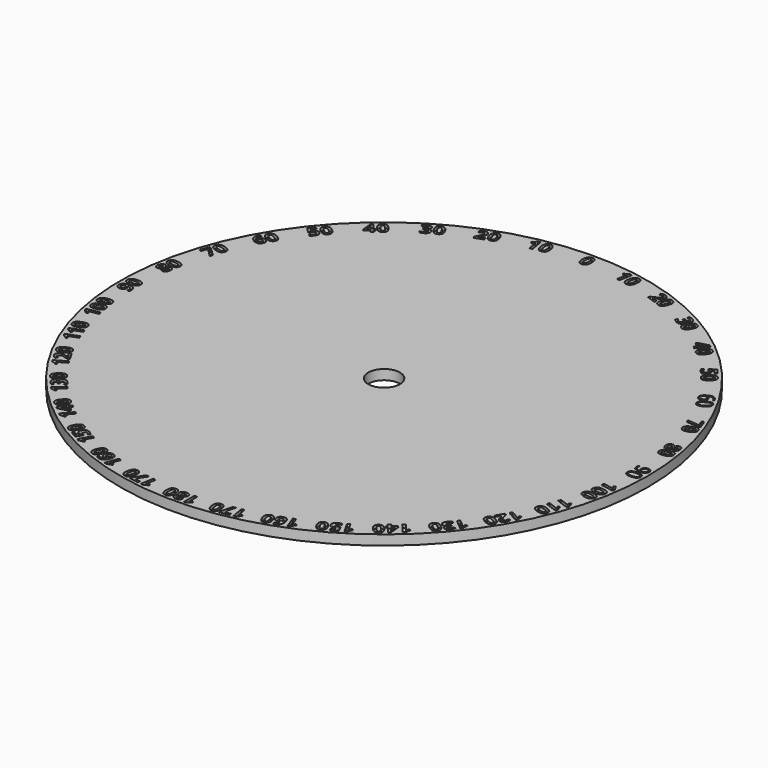
from build123d import *

# Parameters (mm, degrees)
F0_R     = 508
F0_R_2   = 30.48
F1_DEPTH = 19.05
F3_DEPTH = 6.35


with BuildPart() as f1:
    # F0 (on Top) → F1 (new body)
    with BuildSketch(Plane.XY):
        Circle(F0_R)
        Circle(F0_R_2, mode=Mode.SUBTRACT)
    extrude(amount=F1_DEPTH)

    # F2 (on face) → F3 (cut)
    with BuildSketch(Plane.XY.offset(19.05)):
        with BuildLine():
            Line((2.196881654, 476.25), (0, 476.25))
            Line((0, 476.25), (0, 480.240296984))
            add(Edge.make_bspline(
                [(-0.5236545139, 480.1967013889), (-0.2507065353, 480.1967013889), (0, 480.240296984)],
                knots=[0, 0, 0, 0.1465014543, 0.1465014543, 0.1465014543], degree=2))
            add(Edge.make_bspline(
                [(-3.2190972222, 482.203125), (-2.4198350694, 480.1967013889), (-0.5236545139, 480.1967013889)],
                knots=[0, 0, 0, 1, 1, 1], degree=2))
            add(Edge.make_bspline(
                [(-4.018359375, 488.8397569444), (-4.018359375, 484.2095486111), (-3.2190972222, 482.203125)],
                knots=[0, 0, 0, 1, 1, 1], degree=2))
            add(Edge.make_bspline(
                [(-3.2108289931, 495.4984375), (-4.018359375, 493.4754774306), (-4.018359375, 488.8397569444)],
                knots=[0, 0, 0, 1, 1, 1], degree=2))
            add(Edge.make_bspline(
                [(-0.5236545139, 497.5213975694), (-2.4032986111, 497.5213975694), (-3.2108289931, 495.4984375)],
                knots=[0, 0, 0, 1, 1, 1], degree=2))
            add(Edge.make_bspline(
                [(0, 497.4769670954), (-0.2508104364, 497.5213975694), (-0.5236545139, 497.5213975694)],
                knots=[0.8518004728, 0.8518004728, 0.8518004728, 1, 1, 1], degree=2))
            Line((0, 497.4769670954), (0, 501.8196113844))
            add(Edge.make_bspline(
                [(-0.5236545139, 501.8319010417), (-0.2578689632, 501.8319010417), (0, 501.8196113844)],
                knots=[0, 0, 0, 0.0609584109, 0.0609584109, 0.0609584109], degree=2))
            add(Edge.make_bspline(
                [(-7.1547743056, 498.6706814236), (-4.9995225694, 501.8319010417), (-0.5236545139, 501.8319010417)],
                knots=[0, 0, 0, 1, 1, 1], degree=2))
            add(Edge.make_bspline(
                [(-9.3100260417, 488.8397569444), (-9.3100260417, 495.5094618056), (-7.1547743056, 498.6706814236)],
                knots=[0, 0, 0, 1, 1, 1], degree=2))
            add(Edge.make_bspline(
                [(-7.0968967014, 479.176953125), (-9.3100260417, 482.451171875), (-9.3100260417, 488.8397569444)],
                knots=[0, 0, 0, 1, 1, 1], degree=2))
            add(Edge.make_bspline(
                [(-0.5236545139, 475.902734375), (-4.8837673611, 475.902734375), (-7.0968967014, 479.176953125)],
                knots=[0, 0, 0, 1, 1, 1], degree=2))
            add(Edge.make_bspline(
                [(2.196881654, 476.25), (0.9645376578, 475.902734375), (-0.5236545139, 475.902734375)],
                knots=[0.6691374514, 0.6691374514, 0.6691374514, 1, 1, 1], degree=2))
        make_face()
        with BuildLine():
            Line((0, 480.240296984), (0, 476.25))
            Line((0, 476.25), (2.196881654, 476.25))
            add(Edge.make_bspline(
                [(6.1350260417, 479.0749782986), (4.689178, 476.9523110843), (2.196881654, 476.25)],
                knots=[0, 0, 0, 0.6691374514, 0.6691374514, 0.6691374514], degree=2))
            add(Edge.make_bspline(
                [(8.2957899306, 488.8397569444), (8.2957899306, 482.2472222222), (6.1350260417, 479.0749782986)],
                knots=[0, 0, 0, 1, 1, 1], degree=2))
            add(Edge.make_bspline(
                [(6.0661241319, 498.524609375), (8.2957899306, 495.2173177083), (8.2957899306, 488.8397569444)],
                knots=[0, 0, 0, 1, 1, 1], degree=2))
            add(Edge.make_bspline(
                [(0, 501.8196113844), (3.9723752174, 501.6302937971), (6.0661241319, 498.524609375)],
                knots=[0.0609584109, 0.0609584109, 0.0609584109, 1, 1, 1], degree=2))
            Line((0, 501.8196113844), (0, 497.4769670954))
            add(Edge.make_bspline(
                [(2.1552517361, 495.4984375), (1.4415730761, 497.2215958436), (0, 497.4769670954)],
                knots=[0, 0, 0, 0.8518004728, 0.8518004728, 0.8518004728], degree=2))
            add(Edge.make_bspline(
                [(2.9930989583, 488.8397569444), (2.9930989583, 493.4754774306), (2.1552517361, 495.4984375)],
                knots=[0, 0, 0, 1, 1, 1], degree=2))
            add(Edge.make_bspline(
                [(2.1662760417, 482.2279296875), (2.9930989583, 484.2591579861), (2.9930989583, 488.8397569444)],
                knots=[0, 0, 0, 1, 1, 1], degree=2))
            add(Edge.make_bspline(
                [(0, 480.240296984), (1.4605838847, 480.4942792887), (2.1662760417, 482.2279296875)],
                knots=[0.1465014543, 0.1465014543, 0.1465014543, 1, 1, 1], degree=2))
        make_face()
        with BuildLine():
            add(Edge.make_bspline(
                [(89.526722161, 467.8109472992), (87.2204273707, 468.9477492344), (86.1341181067, 471.3812610237)],
                knots=[0.3256694736, 0.3256694736, 0.3256694736, 1, 1, 1], degree=2))
            Line((89.526722161, 467.8109472992), (94.7784430096, 466.8849272185))
            add(Edge.make_bspline(
                [(99.1473104685, 468.9831361527), (97.3548308138, 467.1437859007), (94.7784430096, 466.8849272185)],
                knots=[0, 0, 0, 0.6691374514, 0.6691374514, 0.6691374514], degree=2))
            add(Edge.make_bspline(
                [(102.9708835159, 478.2243531579), (101.8261018752, 471.7319738515), (99.1473104685, 468.9831361527)],
                knots=[0, 0, 0, 1, 1, 1], degree=2))
            add(Edge.make_bspline(
                [(102.4568483263, 488.149248321), (104.0783353205, 484.5050244435), (102.9708835159, 478.2243531579)],
                knots=[0, 0, 0, 1, 1, 1], degree=2))
            add(Edge.make_bspline(
                [(96.5414883962, 492.5505978489), (100.8353613322, 491.7934721986), (102.4568483263, 488.149248321)],
                knots=[0, 0, 0, 1, 1, 1], degree=2))
            add(Edge.make_bspline(
                [(89.4621701884, 490.5888861278), (92.1336188337, 493.3278241802), (96.5414883962, 492.5505978489)],
                knots=[0, 0, 0, 1, 1, 1], degree=2))
            add(Edge.make_bspline(
                [(85.6325394484, 481.2815710178), (86.7907215431, 487.8499480753), (89.4621701884, 490.5888861278)],
                knots=[0, 0, 0, 1, 1, 1], degree=2))
            add(Edge.make_bspline(
                [(86.1341181067, 471.3812610237), (84.5231732932, 474.9900429107), (85.6325394484, 481.2815710178)],
                knots=[0, 0, 0, 1, 1, 1], degree=2))
        make_face()
        with BuildLine():
            add(Edge.make_bspline(
                [(90.843813808, 480.3626827443), (90.0397865687, 475.8028176796), (90.4784943298, 473.6880857352)],
                knots=[0, 0, 0, 1, 1, 1], degree=2))
            add(Edge.make_bspline(
                [(92.7953437331, 486.779976801), (91.6487982226, 484.9279762199), (90.843813808, 480.3626827443)],
                knots=[0, 0, 0, 1, 1, 1], degree=2))
            add(Edge.make_bspline(
                [(95.7929773234, 488.3055806101), (93.9418892436, 488.6319773822), (92.7953437331, 486.779976801)],
                knots=[0, 0, 0, 1, 1, 1], degree=2))
            add(Edge.make_bspline(
                [(98.0799016385, 485.8481666612), (97.6060665278, 487.9858840649), (95.7929773234, 488.3055806101)],
                knots=[0, 0, 0, 1, 1, 1], degree=2))
            add(Edge.make_bspline(
                [(97.7487523346, 479.145155782), (98.5537367492, 483.7104492575), (98.0799016385, 485.8481666612)],
                knots=[0, 0, 0, 1, 1, 1], degree=2))
            add(Edge.make_bspline(
                [(95.7863589617, 472.7773533305), (96.9533396729, 474.6341464144), (97.7487523346, 479.145155782)],
                knots=[0, 0, 0, 1, 1, 1], degree=2))
            add(Edge.make_bspline(
                [(92.7845754031, 471.2440854929), (94.6193782505, 470.9205602466), (95.7863589617, 472.7773533305)],
                knots=[0, 0, 0, 1, 1, 1], degree=2))
            add(Edge.make_bspline(
                [(90.4784943298, 473.6880857352), (90.9172020908, 471.5733537909), (92.7845754031, 471.2440854929)],
                knots=[0, 0, 0, 1, 1, 1], degree=2))
        make_face(mode=Mode.SUBTRACT)
        with BuildLine():
            Line((94.7784430096, 466.8849272185), (89.526722161, 467.8109472992))
            add(Edge.make_bspline(
                [(92.0389358561, 467.0153534864), (90.6405525172, 467.2619261985), (89.526722161, 467.8109472992)],
                knots=[0, 0, 0, 0.3256694736, 0.3256694736, 0.3256694736], degree=2))
            add(Edge.make_bspline(
                [(94.7784430096, 466.8849272185), (93.5045190448, 466.7569316278), (92.0389358561, 467.0153534864)],
                knots=[0.6691374514, 0.6691374514, 0.6691374514, 1, 1, 1], degree=2))
        make_face()
        with BuildLine():
            add(Edge.make_bspline(
                [(169.401128577, 445.1576956885), (167.3272751713, 446.6777109354), (166.6800442734, 449.2628878367)],
                knots=[0.3256694736, 0.3256694736, 0.3256694736, 1, 1, 1], degree=2))
            Line((169.401128577, 445.1576956885), (174.4122622859, 443.3337921785))
            add(Edge.make_bspline(
                [(179.0791069892, 444.6414787317), (176.9944593087, 443.1413331685), (174.4122622859, 443.3337921785)],
                knots=[0, 0, 0, 0.6691374514, 0.6691374514, 0.6691374514], degree=2))
            add(Edge.make_bspline(
                [(184.4493118628, 453.0783443939), (182.1945321922, 446.8833881631), (179.0791069892, 444.6414787317)],
                knots=[0, 0, 0, 1, 1, 1], degree=2))
            add(Edge.make_bspline(
                [(185.6665259814, 462.9417193723), (186.6305661093, 459.0712911823), (184.4493118628, 453.0783443939)],
                knots=[0, 0, 0, 1, 1, 1], degree=2))
            add(Edge.make_bspline(
                [(180.6053199852, 468.3033939832), (184.7024858535, 466.8121475622), (185.6665259814, 462.9417193723)],
                knots=[0, 0, 0, 1, 1, 1], degree=2))
            add(Edge.make_bspline(
                [(173.2929048625, 467.6007957769), (176.3993798017, 469.834231017), (180.6053199852, 468.3033939832)],
                knots=[0, 0, 0, 1, 1, 1], degree=2))
            add(Edge.make_bspline(
                [(167.9052565108, 459.099888096), (170.1864299233, 465.3673605369), (173.2929048625, 467.6007957769)],
                knots=[0, 0, 0, 1, 1, 1], degree=2))
            add(Edge.make_bspline(
                [(166.6800442734, 449.2628878367), (165.7202317297, 453.096581849), (167.9052565108, 459.099888096)],
                knots=[0, 0, 0, 1, 1, 1], degree=2))
        make_face()
        with BuildLine():
            add(Edge.make_bspline(
                [(172.8777966291, 457.2900315043), (171.2941721113, 452.9390589007), (171.3589955673, 450.7802736832)],
                knots=[0, 0, 0, 1, 1, 1], degree=2))
            add(Edge.make_bspline(
                [(175.9140298481, 463.2709528295), (174.4633064142, 461.6461838371), (172.8777966291, 457.2900315043)],
                knots=[0, 0, 0, 1, 1, 1], degree=2))
            add(Edge.make_bspline(
                [(179.1310409698, 464.2528456784), (177.3647532819, 464.895721822), (175.9140298481, 463.2709528295)],
                knots=[0, 0, 0, 1, 1, 1], degree=2))
            add(Edge.make_bspline(
                [(180.9564963118, 461.4356451294), (180.8610705526, 463.6231664059), (179.1310409698, 464.2528456784)],
                knots=[0, 0, 0, 1, 1, 1], degree=2))
            add(Edge.make_bspline(
                [(179.4664122859, 454.8919715202), (181.051922071, 459.248123853), (180.9564963118, 461.4356451294)],
                knots=[0, 0, 0, 1, 1, 1], degree=2))
            add(Edge.make_bspline(
                [(176.4280747863, 448.9616763294), (177.8997551736, 450.5876164803), (179.4664122859, 454.8919715202)],
                knots=[0, 0, 0, 1, 1, 1], degree=2))
            add(Edge.make_bspline(
                [(173.205645899, 447.9729565202), (174.956394399, 447.3357361785), (176.4280747863, 448.9616763294)],
                knots=[0, 0, 0, 1, 1, 1], degree=2))
            add(Edge.make_bspline(
                [(171.3589955673, 450.7802736832), (171.4238190233, 448.6214884656), (173.205645899, 447.9729565202)],
                knots=[0, 0, 0, 1, 1, 1], degree=2))
        make_face(mode=Mode.SUBTRACT)
        with BuildLine():
            Line((174.4122622859, 443.3337921785), (169.401128577, 445.1576956885))
            add(Edge.make_bspline(
                [(171.7370226855, 443.9379474034), (170.4027008338, 444.4236008403), (169.401128577, 445.1576956885)],
                knots=[0, 0, 0, 0.3256694736, 0.3256694736, 0.3256694736], degree=2))
            add(Edge.make_bspline(
                [(174.4122622859, 443.3337921785), (173.1354658876, 443.4289557035), (171.7370226855, 443.9379474034)],
                knots=[0.6691374514, 0.6691374514, 0.6691374514, 1, 1, 1], degree=2))
        make_face()
        with BuildLine():
            add(Edge.make_bspline(
                [(244.1283674224, 408.978552755), (242.3499683874, 410.8355964194), (242.1614816391, 413.4938891407)],
                knots=[0.3256694736, 0.3256694736, 0.3256694736, 1, 1, 1], degree=2))
            Line((244.1283674224, 408.978552755), (248.7466532296, 406.312184201))
            add(Edge.make_bspline(
                [(253.5696754623, 406.7896149789), (251.2562007211, 405.6742552684), (248.7466532296, 406.312184201)],
                knots=[0, 0, 0, 0.6691374514, 0.6691374514, 0.6691374514], degree=2))
            add(Edge.make_bspline(
                [(260.3233412046, 414.1657794041), (257.0270738435, 408.4564768593), (253.5696754623, 406.7896149789)],
                knots=[0, 0, 0, 1, 1, 1], degree=2))
            add(Edge.make_bspline(
                [(263.2348201963, 423.6679405402), (263.5121215865, 419.6889090398), (260.3233412046, 414.1657794041)],
                knots=[0, 0, 0, 1, 1, 1], degree=2))
            add(Edge.make_bspline(
                [(259.1815503171, 429.8270284642), (262.9575188061, 427.6469720405), (263.2348201963, 423.6679405402)],
                knots=[0, 0, 0, 1, 1, 1], degree=2))
            add(Edge.make_bspline(
                [(251.8582223129, 430.4048918638), (255.305334877, 432.0649624919), (259.1815503171, 429.8270284642)],
                knots=[0, 0, 0, 1, 1, 1], degree=2))
            add(Edge.make_bspline(
                [(245.0762573183, 422.9686873902), (248.4111097489, 428.7448212357), (251.8582223129, 430.4048918638)],
                knots=[0, 0, 0, 1, 1, 1], degree=2))
            add(Edge.make_bspline(
                [(242.1614816391, 413.4938891407), (241.8819647836, 417.4360104259), (245.0762573183, 422.9686873902)],
                knots=[0, 0, 0, 1, 1, 1], degree=2))
        make_face()
        with BuildLine():
            add(Edge.make_bspline(
                [(249.65897508, 420.3228540569), (247.3438709133, 416.3129760154), (247.0328404364, 414.175731121)],
                knots=[0, 0, 0, 1, 1, 1], degree=2))
            add(Edge.make_bspline(
                [(253.6876571829, 425.6856753827), (251.976835323, 424.3375057627), (249.65897508, 420.3228540569)],
                knots=[0, 0, 0, 1, 1, 1], degree=2))
            add(Edge.make_bspline(
                [(257.0262985809, 426.0940229541), (255.3984790427, 427.0338450027), (253.6876571829, 425.6856753827)],
                knots=[0, 0, 0, 1, 1, 1], degree=2))
            add(Edge.make_bspline(
                [(258.3348194131, 423.0026350181), (258.6207024689, 425.1734934402), (257.0262985809, 426.0940229541)],
                knots=[0, 0, 0, 1, 1, 1], degree=2))
            add(Edge.make_bspline(
                [(255.7310761142, 416.8171248902), (258.0489363573, 420.831776596), (258.3348194131, 423.0026350181)],
                knots=[0, 0, 0, 1, 1, 1], degree=2))
            add(Edge.make_bspline(
                [(251.7091128355, 411.5045259786), (253.4407766351, 412.8502098278), (255.7310761142, 416.8171248902)],
                knots=[0, 0, 0, 1, 1, 1], degree=2))
            add(Edge.make_bspline(
                [(248.3639504907, 411.0903959489), (249.9774490359, 410.1588421295), (251.7091128355, 411.5045259786)],
                knots=[0, 0, 0, 1, 1, 1], degree=2))
            add(Edge.make_bspline(
                [(247.0328404364, 414.175731121), (246.7218099594, 412.0384862267), (248.3639504907, 411.0903959489)],
                knots=[0, 0, 0, 1, 1, 1], degree=2))
        make_face(mode=Mode.SUBTRACT)
        with BuildLine():
            Line((248.7466532296, 406.312184201), (244.1283674224, 408.978552755))
            add(Edge.make_bspline(
                [(246.2169669837, 407.3717114319), (244.9872493134, 408.0816892598), (244.1283674224, 408.978552755)],
                knots=[0, 0, 0, 0.3256694736, 0.3256694736, 0.3256694736], degree=2))
            add(Edge.make_bspline(
                [(248.7466532296, 406.312184201), (247.5057792101, 406.627615346), (246.2169669837, 407.3717114319)],
                knots=[0.6691374514, 0.6691374514, 0.6691374514, 1, 1, 1], degree=2))
        make_face()
        with BuildLine():
            add(Edge.make_bspline(
                [(311.4378893586, 360.3728034491), (310.0089804492, 362.5104501991), (310.2849649248, 365.1610878611)],
                knots=[0.3256694736, 0.3256694736, 0.3256694736, 1, 1, 1], degree=2))
            Line((311.4378893586, 360.3728034491), (315.5230029867, 356.9449861104))
            add(Edge.make_bspline(
                [(320.355657659, 356.5776546205), (317.8836496163, 355.8809704031), (315.5230029867, 356.9449861104)],
                knots=[0, 0, 0, 0.6691374514, 0.6691374514, 0.6691374514], degree=2))
            add(Edge.make_bspline(
                [(328.2875775539, 362.6689967852), (324.049977918, 357.6188221951), (320.355657659, 356.5776546205)],
                knots=[0, 0, 0, 1, 1, 1], degree=2))
            add(Edge.make_bspline(
                [(332.8048576028, 371.5212257211), (332.3869945929, 367.554491769), (328.2875775539, 362.6689967852)],
                knots=[0, 0, 0, 1, 1, 1], degree=2))
            add(Edge.make_bspline(
                [(329.8826803948, 378.2905861883), (333.2227206127, 375.4879596732), (332.8048576028, 371.5212257211)],
                knots=[0, 0, 0, 1, 1, 1], degree=2))
            add(Edge.make_bspline(
                [(322.7709551247, 380.1313531068), (326.4539665427, 381.167618717), (329.8826803948, 378.2905861883)],
                knots=[0, 0, 0, 1, 1, 1], degree=2))
            add(Edge.make_bspline(
                [(314.8007400618, 373.9857971505), (319.0879437067, 379.0950874966), (322.7709551247, 380.1313531068)],
                knots=[0, 0, 0, 1, 1, 1], degree=2))
            add(Edge.make_bspline(
                [(310.2849649248, 365.1610878611), (310.6942367357, 369.0918570587), (314.8007400618, 373.9857971505)],
                knots=[0, 0, 0, 1, 1, 1], degree=2))
        make_face()
        with BuildLine():
            add(Edge.make_bspline(
                [(318.8543919066, 370.5843793826), (315.8781513597, 367.0374340184), (315.2007174534, 364.9866685518)],
                knots=[0, 0, 0, 1, 1, 1], degree=2))
            add(Edge.make_bspline(
                [(323.7531134263, 375.1661540967), (321.834175597, 374.1355473009), (318.8543919066, 370.5843793826)],
                knots=[0, 0, 0, 1, 1, 1], degree=2))
            add(Edge.make_bspline(
                [(327.1119421713, 374.9885489563), (325.6720512556, 376.1967608926), (323.7531134263, 375.1661540967)],
                knots=[0, 0, 0, 1, 1, 1], degree=2))
            add(Edge.make_bspline(
                [(327.8637697502, 371.7169038915), (328.522275209, 373.8051390246), (327.1119421713, 374.9885489563)],
                knots=[0, 0, 0, 1, 1, 1], degree=2))
            add(Edge.make_bspline(
                [(324.225480601, 366.0775008401), (327.2052642915, 369.6286687584), (327.8637697502, 371.7169038915)],
                knots=[0, 0, 0, 1, 1, 1], degree=2))
            add(Edge.make_bspline(
                [(319.3420968621, 361.5440188373), (321.2811283456, 362.5685584619), (324.225480601, 366.0775008401)],
                knots=[0, 0, 0, 1, 1, 1], degree=2))
            add(Edge.make_bspline(
                [(315.9758421249, 361.7170617185), (317.4030653786, 360.5194792127), (319.3420968621, 361.5440188373)],
                knots=[0, 0, 0, 1, 1, 1], degree=2))
            add(Edge.make_bspline(
                [(315.2007174534, 364.9866685518), (314.5232835471, 362.9359030853), (315.9758421249, 361.7170617185)],
                knots=[0, 0, 0, 1, 1, 1], degree=2))
        make_face(mode=Mode.SUBTRACT)
        with BuildLine():
            Line((315.5230029867, 356.9449861104), (311.4378893586, 360.3728034491))
            add(Edge.make_bspline(
                [(313.2157333319, 358.4276921486), (312.1279841922, 359.3404220505), (311.4378893586, 360.3728034491)],
                knots=[0, 0, 0, 0.3256694736, 0.3256694736, 0.3256694736], degree=2))
            add(Edge.make_bspline(
                [(315.5230029867, 356.9449861104), (314.3557546754, 357.4711006597), (313.2157333319, 358.4276921486)],
                knots=[0.6691374514, 0.6691374514, 0.6691374514, 1, 1, 1], degree=2))
        make_face()
        with BuildLine():
            add(Edge.make_bspline(
                [(369.2845286217, 300.8173088679), (368.248526512, 303.1706073887), (368.980596563, 305.7330517074)],
                knots=[0.3256694736, 0.3256694736, 0.3256694736, 1, 1, 1], degree=2))
            Line((369.2845286217, 300.8173088679), (372.7123459604, 296.7321952397))
            add(Edge.make_bspline(
                [(377.4077953055, 295.5312626634), (374.8523646747, 295.2744223365), (372.7123459604, 296.7321952397)],
                knots=[0, 0, 0, 0.6691374514, 0.6691374514, 0.6691374514], degree=2))
            add(Edge.make_bspline(
                [(386.2769619807, 300.1527002183), (381.2267873906, 295.9151005824), (377.4077953055, 295.5312626634)],
                knots=[0, 0, 0, 1, 1, 1], degree=2))
            add(Edge.make_bspline(
                [(392.2627878184, 308.0860264573), (391.1624569645, 304.2521172573), (386.2769619807, 300.1527002183)],
                knots=[0, 0, 0, 1, 1, 1], degree=2))
            add(Edge.make_bspline(
                [(390.5604921573, 315.2599758753), (393.3631186724, 311.9199356573), (392.2627878184, 308.0860264573)],
                knots=[0, 0, 0, 1, 1, 1], degree=2))
            add(Edge.make_bspline(
                [(383.876455795, 318.3077155414), (387.6834596286, 318.6886897274), (390.5604921573, 315.2599758753)],
                knots=[0, 0, 0, 1, 1, 1], degree=2))
            add(Edge.make_bspline(
                [(374.9601616153, 313.6395377104), (380.0694519614, 317.9267413554), (383.876455795, 318.3077155414)],
                knots=[0, 0, 0, 1, 1, 1], degree=2))
            add(Edge.make_bspline(
                [(368.980596563, 305.7330517074), (370.0662215235, 309.5330343843), (374.9601616153, 313.6395377104)],
                knots=[0, 0, 0, 1, 1, 1], degree=2))
        make_face()
        with BuildLine():
            add(Edge.make_bspline(
                [(378.3615793832, 309.5858858655), (374.814634019, 306.6096453186), (373.7913801699, 304.7076707509)],
                knots=[0, 0, 0, 1, 1, 1], degree=2))
            add(Edge.make_bspline(
                [(383.9814951453, 313.2473990618), (381.9127473015, 312.565669556), (378.3615793832, 309.5858858655)],
                knots=[0, 0, 0, 1, 1, 1], degree=2))
            add(Edge.make_bspline(
                [(387.2584549254, 312.4892376518), (386.0502429891, 313.9291285676), (383.9814951453, 313.2473990618)],
                knots=[0, 0, 0, 1, 1, 1], degree=2))
            add(Edge.make_bspline(
                [(387.4307453506, 309.1367427379), (388.4418648572, 311.0789046142), (387.2584549254, 312.4892376518)],
                knots=[0, 0, 0, 1, 1, 1], degree=2))
            add(Edge.make_bspline(
                [(382.8684579257, 304.2147971711), (386.419625844, 307.1945808616), (387.4307453506, 309.1367427379)],
                knots=[0, 0, 0, 1, 1, 1], degree=2))
            add(Edge.make_bspline(
                [(377.2720328705, 300.5981796337), (379.3595155475, 301.2704449158), (382.8684579257, 304.2147971711)],
                knots=[0, 0, 0, 1, 1, 1], degree=2))
            add(Edge.make_bspline(
                [(373.9869676876, 301.3531376054), (375.1845501934, 299.9259143517), (377.2720328705, 300.5981796337)],
                knots=[0, 0, 0, 1, 1, 1], degree=2))
            add(Edge.make_bspline(
                [(373.7913801699, 304.7076707509), (372.7681263207, 302.8056961831), (373.9869676876, 301.3531376054)],
                knots=[0, 0, 0, 1, 1, 1], degree=2))
        make_face(mode=Mode.SUBTRACT)
        with BuildLine():
            Line((372.7123459604, 296.7321952397), (369.2845286217, 300.8173088679))
            add(Edge.make_bspline(
                [(370.6975981176, 298.5930288125), (369.7848682157, 299.6807779522), (369.2845286217, 300.8173088679)],
                knots=[0, 0, 0, 0.3256694736, 0.3256694736, 0.3256694736], degree=2))
            add(Edge.make_bspline(
                [(372.7123459604, 296.7321952397), (371.6541896064, 297.453007469), (370.6975981176, 298.5930288125)],
                knots=[0.6691374514, 0.6691374514, 0.6691374514, 1, 1, 1], degree=2))
        make_face()
        with BuildLine():
            add(Edge.make_bspline(
                [(416.1249982319, 231.7503607628), (415.5919288992, 234.1198217625), (416.8061258385, 236.4741287668)],
                knots=[0.3244428423, 0.3244428423, 0.3244428423, 1, 1, 1], degree=2))
            Line((416.1249982319, 231.7503607628), (418.6149160201, 227.4376966471))
            add(Edge.make_bspline(
                [(422.9790514823, 225.6279676427), (420.4134458649, 225.7435239542), (418.6149160201, 227.4376966471)],
                knots=[0, 0, 0, 0.6716946069, 0.6716946069, 0.6716946069], degree=2))
            add(Edge.make_bspline(
                [(432.4554450545, 228.7218811836), (426.7986528174, 225.4559306628), (422.9790514823, 225.6279676427)],
                knots=[0, 0, 0, 1, 1, 1], degree=2))
            add(Edge.make_bspline(
                [(439.7288043296, 235.3780030302), (437.9117433895, 231.8720764961), (432.4554450545, 228.7218811836)],
                knots=[0, 0, 0, 1, 1, 1], degree=2))
            add(Edge.make_bspline(
                [(439.4953444364, 242.4355358295), (441.5458652697, 238.8839295642), (439.7288043296, 235.3780030302)],
                knots=[0, 0, 0, 1, 1, 1], degree=2))
            add(Edge.make_bspline(
                [(433.6083889935, 246.2544809946), (437.395214228, 246.0730680529), (439.4953444364, 242.4355358295)],
                knots=[0, 0, 0, 1, 1, 1], degree=2))
            add(Edge.make_bspline(
                [(424.1265822072, 243.1478948043), (429.821563759, 246.4358939362), (433.6083889935, 246.2544809946)],
                knots=[0, 0, 0, 1, 1, 1], degree=2))
            add(Edge.make_bspline(
                [(416.8061258385, 236.4741287668), (418.6034525715, 239.9591144224), (424.1265822072, 243.1478948043)],
                knots=[0, 0, 0, 1, 1, 1], degree=2))
        make_face()
        with BuildLine():
            add(Edge.make_bspline(
                [(425.5735223114, 240.6417210284), (420.8141789693, 237.8939128687), (419.28846161, 235.5204738251)],
                knots=[0, 0, 0, 1, 1, 1], degree=2))
            add(Edge.make_bspline(
                [(433.134475014, 243.5144733911), (430.3328656535, 243.3895291881), (425.5735223114, 240.6417210284)],
                knots=[0, 0, 0, 1, 1, 1], degree=2))
            add(Edge.make_bspline(
                [(437.3471954856, 241.1953014545), (435.9360843745, 243.6394175941), (433.134475014, 243.5144733911)],
                knots=[0, 0, 0, 1, 1, 1], degree=2))
            add(Edge.make_bspline(
                [(437.2320486264, 236.3456097206), (438.7775991314, 238.7177696646), (437.3471954856, 241.1953014545)],
                knots=[0, 0, 0, 1, 1, 1], degree=2))
            add(Edge.make_bspline(
                [(430.9892124156, 231.2614706099), (435.6864981213, 233.9734497766), (437.2320486264, 236.3456097206)],
                knots=[0, 0, 0, 1, 1, 1], degree=2))
            add(Edge.make_bspline(
                [(423.4457060266, 228.3860611095), (426.2871530455, 228.5467353669), (430.9892124156, 231.2614706099)],
                knots=[0, 0, 0, 1, 1, 1], degree=2))
            add(Edge.make_bspline(
                [(419.1738553619, 230.702918642), (420.6042590077, 228.2253868521), (423.4457060266, 228.3860611095)],
                knots=[0, 0, 0, 1, 1, 1], degree=2))
            add(Edge.make_bspline(
                [(419.28846161, 235.5204738251), (417.7627442508, 233.1470347816), (419.1738553619, 230.702918642)],
                knots=[0, 0, 0, 1, 1, 1], degree=2))
        make_face(mode=Mode.SUBTRACT)
        with BuildLine():
            Line((418.6149160201, 227.4376966471), (416.1249982319, 231.7503607628))
            add(Edge.make_bspline(
                [(417.0400274041, 229.4709524962), (416.3810099216, 230.6124042589), (416.1249982319, 231.7503607628)],
                knots=[0, 0, 0, 0.3244428423, 0.3244428423, 0.3244428423], degree=2))
            add(Edge.make_bspline(
                [(418.6149160201, 227.4376966471), (417.7358453209, 228.2657605115), (417.0400274041, 229.4709524962)],
                knots=[0.6716946069, 0.6716946069, 0.6716946069, 1, 1, 1], degree=2))
        make_face()
        with BuildLine():
            add(Edge.make_bspline(
                [(449.8995256101, 156.3730579407), (449.7308775699, 158.9387687852), (451.2952059678, 161.0962960989)],
                knots=[0.3256694736, 0.3256694736, 0.3256694736, 1, 1, 1], degree=2))
            Line((449.8995256101, 156.3730579407), (451.72342912, 151.3619242318))
            add(Edge.make_bspline(
                [(455.724965089, 148.6274784937), (453.2358012169, 149.2601362844), (451.72342912, 151.3619242318)],
                knots=[0, 0, 0, 0.6691374514, 0.6691374514, 0.6691374514], degree=2))
            add(Edge.make_bspline(
                [(465.6398803011, 149.936775604), (459.4449240703, 147.6819959335), (455.724965089, 148.6274784937)],
                knots=[0, 0, 0, 1, 1, 1], degree=2))
            add(Edge.make_bspline(
                [(473.9780740475, 155.3443907182), (471.6328270895, 152.1180298506), (465.6398803011, 149.936775604)],
                knots=[0, 0, 0, 1, 1, 1], degree=2))
            add(Edge.make_bspline(
                [(474.8320745845, 162.6679174542), (476.3233210054, 158.5707515858), (473.9780740475, 155.3443907182)],
                knots=[0, 0, 0, 1, 1, 1], degree=2))
            add(Edge.make_bspline(
                [(469.5935232952, 167.8179310031), (473.3012375506, 166.8738576376), (474.8320745845, 162.6679174542)],
                knots=[0, 0, 0, 1, 1, 1], degree=2))
            add(Edge.make_bspline(
                [(459.6183365989, 166.4808309561), (465.8858090397, 168.7620043686), (469.5935232952, 167.8179310031)],
                knots=[0, 0, 0, 1, 1, 1], degree=2))
            add(Edge.make_bspline(
                [(451.2952059678, 161.0962960989), (453.6150303519, 164.295806175), (459.6183365989, 166.4808309561)],
                knots=[0, 0, 0, 1, 1, 1], degree=2))
        make_face()
        with BuildLine():
            add(Edge.make_bspline(
                [(461.4281931907, 161.5082908377), (457.0772205871, 159.9246663199), (455.4651628816, 158.4873682819)],
                knots=[0, 0, 0, 1, 1, 1], degree=2))
            add(Edge.make_bspline(
                [(467.9614978299, 163.0268633747), (465.7843455235, 163.0938006228), (461.4281931907, 161.5082908377)],
                knots=[0, 0, 0, 1, 1, 1], degree=2))
            add(Edge.make_bspline(
                [(470.7815262798, 161.1936384388), (470.1386501362, 162.9599261267), (467.9614978299, 163.0268633747)],
                knots=[0, 0, 0, 1, 1, 1], degree=2))
            add(Edge.make_bspline(
                [(469.7968055299, 157.984396911), (471.4112055523, 159.463608856), (470.7815262798, 161.1936384388)],
                knots=[0, 0, 0, 1, 1, 1], degree=2))
            add(Edge.make_bspline(
                [(463.8262531747, 154.919675181), (468.1824055076, 156.505184966), (469.7968055299, 157.984396911)],
                knots=[0, 0, 0, 1, 1, 1], degree=2))
            add(Edge.make_bspline(
                [(457.330377799, 153.4352564684), (459.5218981348, 153.3530180687), (463.8262531747, 154.919675181)],
                knots=[0, 0, 0, 1, 1, 1], degree=2))
            add(Edge.make_bspline(
                [(454.5016371215, 155.268243368), (455.1388574632, 153.517494868), (457.330377799, 153.4352564684)],
                knots=[0, 0, 0, 1, 1, 1], degree=2))
            add(Edge.make_bspline(
                [(455.4651628816, 158.4873682819), (453.8531051762, 157.0500702438), (454.5016371215, 155.268243368)],
                knots=[0, 0, 0, 1, 1, 1], degree=2))
        make_face(mode=Mode.SUBTRACT)
        with BuildLine():
            Line((451.72342912, 151.3619242318), (449.8995256101, 156.3730579407))
            add(Edge.make_bspline(
                [(450.4666280047, 153.7996201545), (449.9809745677, 155.1339420063), (449.8995256101, 156.3730579407)],
                knots=[0, 0, 0, 0.3256694736, 0.3256694736, 0.3256694736], degree=2))
            add(Edge.make_bspline(
                [(451.72342912, 151.3619242318), (450.9756197046, 152.4011769524), (450.4666280047, 153.7996201545)],
                knots=[0.6691374514, 0.6691374514, 0.6691374514, 1, 1, 1], degree=2))
        make_face()
        with BuildLine():
            add(Edge.make_bspline(
                [(470.2184374449, 75.8731670668), (470.49788256, 78.4291844233), (472.4130959808, 80.2822912736)],
                knots=[0.3256694736, 0.3256694736, 0.3256694736, 1, 1, 1], degree=2))
            Line((470.2184374449, 75.8731670668), (471.1444575257, 70.6214462181))
            add(Edge.make_bspline(
                [(474.6103696525, 67.2336834262), (472.2688816452, 68.2889684938), (471.1444575257, 70.6214462181)],
                knots=[0, 0, 0, 0.6691374514, 0.6691374514, 0.6691374514], degree=2))
            add(Edge.make_bspline(
                [(484.6020120811, 66.8013824132), (478.1096327746, 65.6566007725), (474.6103696525, 67.2336834262)],
                knots=[0, 0, 0, 1, 1, 1], degree=2))
            add(Edge.make_bspline(
                [(493.7525524387, 70.6789315538), (490.8826833667, 67.9088342178), (484.6020120811, 66.8013824132)],
                knots=[0, 0, 0, 1, 1, 1], degree=2))
            add(Edge.make_bspline(
                [(495.8652958605, 77.7429018258), (496.6224215108, 73.4490288899), (493.7525524387, 70.6789315538)],
                knots=[0, 0, 0, 1, 1, 1], degree=2))
            add(Edge.make_bspline(
                [(491.6006204039, 83.7243399819), (495.0880695291, 82.1507713884), (495.8652958605, 77.7429018258)],
                knots=[0, 0, 0, 1, 1, 1], degree=2))
            add(Edge.make_bspline(
                [(481.5447942212, 84.1397264807), (488.1131712787, 85.2979085754), (491.6006204039, 83.7243399819)],
                knots=[0, 0, 0, 1, 1, 1], degree=2))
            add(Edge.make_bspline(
                [(472.4130959808, 80.2822912736), (475.253266114, 83.0303603256), (481.5447942212, 84.1397264807)],
                knots=[0, 0, 0, 1, 1, 1], degree=2))
        make_face()
        with BuildLine():
            add(Edge.make_bspline(
                [(482.4636824947, 78.928452121), (477.9038174299, 78.1244248817), (476.0666663182, 76.9888935133)],
                knots=[0, 0, 0, 1, 1, 1], degree=2))
            add(Edge.make_bspline(
                [(489.1614289098, 79.2894576843), (487.0289759702, 79.7334365356), (482.4636824947, 78.928452121)],
                knots=[0, 0, 0, 1, 1, 1], degree=2))
            add(Edge.make_bspline(
                [(491.6202786216, 76.994390753), (491.2938818495, 78.8454788329), (489.1614289098, 79.2894576843)],
                knots=[0, 0, 0, 1, 1, 1], degree=2))
            add(Edge.make_bspline(
                [(490.0932390497, 74.0048997789), (491.9399751668, 75.1813015487), (491.6202786216, 76.994390753)],
                knots=[0, 0, 0, 1, 1, 1], degree=2))
            add(Edge.make_bspline(
                [(483.681209457, 72.0235135945), (488.2465029325, 72.828498009), (490.0932390497, 74.0048997789)],
                knots=[0, 0, 0, 1, 1, 1], degree=2))
            add(Edge.make_bspline(
                [(477.0262544201, 71.6896434589), (479.1702000894, 71.2281009327), (483.681209457, 72.0235135945)],
                knots=[0, 0, 0, 1, 1, 1], degree=2))
            add(Edge.make_bspline(
                [(474.5587835044, 73.9859888326), (474.8823087507, 72.1511859852), (477.0262544201, 71.6896434589)],
                knots=[0, 0, 0, 1, 1, 1], degree=2))
            add(Edge.make_bspline(
                [(476.0666663182, 76.9888935133), (474.2295152064, 75.8533621449), (474.5587835044, 73.9859888326)],
                knots=[0, 0, 0, 1, 1, 1], degree=2))
        make_face(mode=Mode.SUBTRACT)
        with BuildLine():
            Line((471.1444575257, 70.6214462181), (470.2184374449, 75.8731670668))
            add(Edge.make_bspline(
                [(470.330051498, 73.2403492857), (470.083478786, 74.6387326246), (470.2184374449, 75.8731670668)],
                knots=[0, 0, 0, 0.3256694736, 0.3256694736, 0.3256694736], degree=2))
            add(Edge.make_bspline(
                [(471.1444575257, 70.6214462181), (470.5884733566, 71.774766097), (470.330051498, 73.2403492857)],
                knots=[0.6691374514, 0.6691374514, 0.6691374514, 1, 1, 1], degree=2))
        make_face()
        with BuildLine():
            add(Edge.make_bspline(
                [(476.25, -7.3607993592), (476.9730789157, -5.0422512738), (479.2017578125, -3.6104600694)],
                knots=[0.3244428423, 0.3244428423, 0.3244428423, 1, 1, 1], degree=2))
            Line((476.25, -7.3607993592), (476.25, -12.3406349355))
            add(Edge.make_bspline(
                [(479.1245876736, -16.0899739583), (476.9604861887, -14.7070964483), (476.25, -12.3406349355)],
                knots=[0, 0, 0, 0.6716946069, 0.6716946069, 0.6716946069], degree=2))
            add(Edge.make_bspline(
                [(488.8783420139, -18.1487630208), (482.3464409722, -18.1487630208), (479.1245876736, -16.0899739583)],
                knots=[0, 0, 0, 1, 1, 1], degree=2))
            add(Edge.make_bspline(
                [(498.5053168403, -16.0210720486), (495.1787326389, -18.1487630208), (488.8783420139, -18.1487630208)],
                knots=[0, 0, 0, 1, 1, 1], degree=2))
            add(Edge.make_bspline(
                [(501.8319010417, -9.7923394097), (501.8319010417, -13.8933810764), (498.5053168403, -16.0210720486)],
                knots=[0, 0, 0, 1, 1, 1], degree=2))
            add(Edge.make_bspline(
                [(498.6431206597, -3.5415581597), (501.8319010417, -5.5920789931), (501.8319010417, -9.7923394097)],
                knots=[0, 0, 0, 1, 1, 1], degree=2))
            add(Edge.make_bspline(
                [(488.8783420139, -1.4910373264), (495.4543402778, -1.4910373264), (498.6431206597, -3.5415581597)],
                knots=[0, 0, 0, 1, 1, 1], degree=2))
            add(Edge.make_bspline(
                [(479.2017578125, -3.6104600694), (482.50078125, -1.4910373264), (488.8783420139, -1.4910373264)],
                knots=[0, 0, 0, 1, 1, 1], degree=2))
        make_face()
        with BuildLine():
            add(Edge.make_bspline(
                [(488.8783420139, -4.3849175347), (483.3827256944, -4.3849175347), (480.8746961806, -5.6775173611)],
                knots=[0, 0, 0, 1, 1, 1], degree=2))
            add(Edge.make_bspline(
                [(496.8626953125, -5.6775173611), (494.3739583333, -4.3849175347), (488.8783420139, -4.3849175347)],
                knots=[0, 0, 0, 1, 1, 1], degree=2))
            add(Edge.make_bspline(
                [(499.3514322917, -9.7923394097), (499.3514322917, -6.9701171875), (496.8626953125, -5.6775173611)],
                knots=[0, 0, 0, 1, 1, 1], degree=2))
            add(Edge.make_bspline(
                [(496.8268663194, -13.9347222222), (499.3514322917, -12.6531467014), (499.3514322917, -9.7923394097)],
                knots=[0, 0, 0, 1, 1, 1], degree=2))
            add(Edge.make_bspline(
                [(488.8783420139, -15.2162977431), (494.3023003472, -15.2162977431), (496.8268663194, -13.9347222222)],
                knots=[0, 0, 0, 1, 1, 1], degree=2))
            add(Edge.make_bspline(
                [(480.9077690972, -13.9347222222), (483.4488715278, -15.2162977431), (488.8783420139, -15.2162977431)],
                knots=[0, 0, 0, 1, 1, 1], degree=2))
            add(Edge.make_bspline(
                [(478.3666666667, -9.7923394097), (478.3666666667, -12.6531467014), (480.9077690972, -13.9347222222)],
                knots=[0, 0, 0, 1, 1, 1], degree=2))
            add(Edge.make_bspline(
                [(480.8746961806, -5.6775173611), (478.3666666667, -6.9701171875), (478.3666666667, -9.7923394097)],
                knots=[0, 0, 0, 1, 1, 1], degree=2))
        make_face(mode=Mode.SUBTRACT)
        with BuildLine():
            Line((476.25, -12.3406349355), (476.25, -7.3607993592))
            add(Edge.make_bspline(
                [(475.902734375, -9.7923394097), (475.902734375, -8.4743044448), (476.25, -7.3607993592)],
                knots=[0, 0, 0, 0.3244428423, 0.3244428423, 0.3244428423], degree=2))
            add(Edge.make_bspline(
                [(476.25, -12.3406349355), (475.902734375, -11.1839752433), (475.902734375, -9.7923394097)],
                knots=[0.6716946069, 0.6716946069, 0.6716946069, 1, 1, 1], degree=2))
        make_face()
        with BuildLine():
            Line((468.6332078763, -84.8634506992), (469.0146923721, -82.6999446139))
            Line((469.0146923721, -82.6999446139), (472.9443677787, -83.3928524135))
            add(Edge.make_bspline(
                [(472.9923661507, -82.8695830927), (472.9449692316, -83.1383843782), (472.9443677787, -83.3928524135)],
                knots=[0, 0, 0, 0.1465014543, 0.1465014543, 0.1465014543], degree=2))
            add(Edge.make_bspline(
                [(475.4363663931, -80.5635020194), (473.3216344487, -81.0022097805), (472.9923661507, -82.8695830927)],
                knots=[0, 0, 0, 1, 1, 1], degree=2))
            add(Edge.make_bspline(
                [(482.1109634022, -80.9288214977), (477.5510983374, -80.1247942584), (475.4363663931, -80.5635020194)],
                knots=[0, 0, 0, 1, 1, 1], degree=2))
            add(Edge.make_bspline(
                [(488.5282574589, -82.8803514227), (486.6762568777, -81.7338059122), (482.1109634022, -80.9288214977)],
                knots=[0, 0, 0, 1, 1, 1], degree=2))
            add(Edge.make_bspline(
                [(490.0538612679, -85.8779850131), (490.3802580401, -84.0268969332), (488.5282574589, -82.8803514227)],
                knots=[0, 0, 0, 1, 1, 1], degree=2))
            add(Edge.make_bspline(
                [(489.9191741406, -86.3859687674), (490.0064823911, -86.1466839759), (490.0538612679, -85.8779850131)],
                knots=[0.8518004728, 0.8518004728, 0.8518004728, 1, 1, 1], degree=2))
            Line((489.9191741406, -86.3859687674), (494.1958439049, -87.1400610344))
            add(Edge.make_bspline(
                [(494.2988785068, -86.6264960858), (494.2527253302, -86.8882437568), (494.1958439049, -87.1400610344)],
                knots=[0, 0, 0, 0.0609584109, 0.0609584109, 0.0609584109], degree=2))
            add(Edge.make_bspline(
                [(492.3371667856, -79.547177878), (495.0761048381, -82.2186265233), (494.2988785068, -86.6264960858)],
                knots=[0, 0, 0, 1, 1, 1], degree=2))
            add(Edge.make_bspline(
                [(483.0298516757, -75.717547138), (489.5982287332, -76.8757292327), (492.3371667856, -79.547177878)],
                knots=[0, 0, 0, 1, 1, 1], degree=2))
            add(Edge.make_bspline(
                [(473.1295416816, -76.2191257963), (476.7383235685, -74.6081809828), (483.0298516757, -75.717547138)],
                knots=[0, 0, 0, 1, 1, 1], degree=2))
            add(Edge.make_bspline(
                [(468.7636341443, -82.1239435458), (469.5207597946, -77.8300706098), (473.1295416816, -76.2191257963)],
                knots=[0, 0, 0, 1, 1, 1], degree=2))
            add(Edge.make_bspline(
                [(468.6332078763, -84.8634506992), (468.5052122856, -83.5895267344), (468.7636341443, -82.1239435458)],
                knots=[0.6691374514, 0.6691374514, 0.6691374514, 1, 1, 1], degree=2))
        make_face()
        with BuildLine():
            Line((472.9443677787, -83.3928524135), (469.0146923721, -82.6999446139))
            Line((469.0146923721, -82.6999446139), (468.6332078763, -84.8634506992))
            add(Edge.make_bspline(
                [(470.7314168106, -89.2323181581), (468.8920665585, -87.4398385035), (468.6332078763, -84.8634506992)],
                knots=[0, 0, 0, 0.6691374514, 0.6691374514, 0.6691374514], degree=2))
            add(Edge.make_bspline(
                [(479.9726338157, -93.0558912055), (473.4802545093, -91.9111095648), (470.7314168106, -89.2323181581)],
                knots=[0, 0, 0, 1, 1, 1], degree=2))
            add(Edge.make_bspline(
                [(489.8975289789, -92.541856016), (486.2533051013, -94.1633430101), (479.9726338157, -93.0558912055)],
                knots=[0, 0, 0, 1, 1, 1], degree=2))
            add(Edge.make_bspline(
                [(494.1958439049, -87.1400610344), (493.3196067597, -91.0192122923), (489.8975289789, -92.541856016)],
                knots=[0.0609584109, 0.0609584109, 0.0609584109, 1, 1, 1], degree=2))
            Line((494.1958439049, -87.1400610344), (489.9191741406, -86.3859687674))
            add(Edge.make_bspline(
                [(487.596447319, -88.1649093281), (489.4173560142, -87.7612963568), (489.9191741406, -86.3859687674)],
                knots=[0, 0, 0, 0.8518004728, 0.8518004728, 0.8518004728], degree=2))
            add(Edge.make_bspline(
                [(480.8934364398, -87.8337600242), (485.4587299153, -88.6387444388), (487.596447319, -88.1649093281)],
                knots=[0, 0, 0, 1, 1, 1], degree=2))
            add(Edge.make_bspline(
                [(474.5256339883, -85.8713666513), (476.3824270722, -87.0383473625), (480.8934364398, -87.8337600242)],
                knots=[0, 0, 0, 1, 1, 1], degree=2))
            add(Edge.make_bspline(
                [(472.9443677787, -83.3928524135), (472.9408637916, -84.8753503115), (474.5256339883, -85.8713666513)],
                knots=[0.1465014543, 0.1465014543, 0.1465014543, 1, 1, 1], degree=2))
        make_face()
        with BuildLine():
            add(Edge.make_bspline(
                [(466.0626666414, -99.4417144714), (467.1994685765, -97.1354196811), (469.6329803659, -96.0491104171)],
                knots=[0.3256694736, 0.3256694736, 0.3256694736, 1, 1, 1], degree=2))
            Line((466.0626666414, -99.4417144714), (465.1366465606, -104.69343532))
            add(Edge.make_bspline(
                [(467.2348554949, -109.0623027789), (465.3955052428, -107.2698231242), (465.1366465606, -104.69343532)],
                knots=[0, 0, 0, 0.6691374514, 0.6691374514, 0.6691374514], degree=2))
            add(Edge.make_bspline(
                [(476.4760725001, -112.8858758263), (469.9836931936, -111.7410941856), (467.2348554949, -109.0623027789)],
                knots=[0, 0, 0, 1, 1, 1], degree=2))
            add(Edge.make_bspline(
                [(486.4009676632, -112.3718406367), (482.7567437857, -113.9933276309), (476.4760725001, -112.8858758263)],
                knots=[0, 0, 0, 1, 1, 1], degree=2))
            add(Edge.make_bspline(
                [(490.8023171911, -106.4564807066), (490.0451915407, -110.7503536426), (486.4009676632, -112.3718406367)],
                knots=[0, 0, 0, 1, 1, 1], degree=2))
            add(Edge.make_bspline(
                [(488.84060547, -99.3771624988), (491.5795435224, -102.048611144), (490.8023171911, -106.4564807066)],
                knots=[0, 0, 0, 1, 1, 1], degree=2))
            add(Edge.make_bspline(
                [(479.53329036, -95.5475317587), (486.1016674175, -96.7057138535), (488.84060547, -99.3771624988)],
                knots=[0, 0, 0, 1, 1, 1], degree=2))
            add(Edge.make_bspline(
                [(469.6329803659, -96.0491104171), (473.2417622528, -94.4381656036), (479.53329036, -95.5475317587)],
                knots=[0, 0, 0, 1, 1, 1], degree=2))
        make_face()
        with BuildLine():
            add(Edge.make_bspline(
                [(478.6144020865, -100.7588061184), (474.0545370218, -99.9547788791), (471.9398050774, -100.3934866402)],
                knots=[0, 0, 0, 1, 1, 1], degree=2))
            add(Edge.make_bspline(
                [(485.0316961432, -102.7103360435), (483.179695562, -101.563790533), (478.6144020865, -100.7588061184)],
                knots=[0, 0, 0, 1, 1, 1], degree=2))
            add(Edge.make_bspline(
                [(486.5572999522, -105.7079696338), (486.8836967244, -103.856881554), (485.0316961432, -102.7103360435)],
                knots=[0, 0, 0, 1, 1, 1], degree=2))
            add(Edge.make_bspline(
                [(484.0998860034, -107.9948939489), (486.2376034071, -107.5210588381), (486.5572999522, -105.7079696338)],
                knots=[0, 0, 0, 1, 1, 1], degree=2))
            add(Edge.make_bspline(
                [(477.3968751241, -107.663744645), (481.9621685996, -108.4687290596), (484.0998860034, -107.9948939489)],
                knots=[0, 0, 0, 1, 1, 1], degree=2))
            add(Edge.make_bspline(
                [(471.0290726726, -105.7013512721), (472.8858657565, -106.8683319833), (477.3968751241, -107.663744645)],
                knots=[0, 0, 0, 1, 1, 1], degree=2))
            add(Edge.make_bspline(
                [(469.4958048351, -102.6995677135), (469.1722795888, -104.5343705609), (471.0290726726, -105.7013512721)],
                knots=[0, 0, 0, 1, 1, 1], degree=2))
            add(Edge.make_bspline(
                [(471.9398050774, -100.3934866402), (469.8250731331, -100.8321944012), (469.4958048351, -102.6995677135)],
                knots=[0, 0, 0, 1, 1, 1], degree=2))
        make_face(mode=Mode.SUBTRACT)
        with BuildLine():
            Line((465.1366465606, -104.69343532), (466.0626666414, -99.4417144714))
            add(Edge.make_bspline(
                [(465.2670728286, -101.9539281665), (465.5136455406, -100.5555448276), (466.0626666414, -99.4417144714)],
                knots=[0, 0, 0, 0.3256694736, 0.3256694736, 0.3256694736], degree=2))
            add(Edge.make_bspline(
                [(465.1366465606, -104.69343532), (465.00865097, -103.4195113552), (465.2670728286, -101.9539281665)],
                knots=[0.6691374514, 0.6691374514, 0.6691374514, 1, 1, 1], degree=2))
        make_face()
        with BuildLine():
            Line((447.9848453318, -161.6335987707), (447.5286106493, -162.8870932588))
            Line((447.5286106493, -162.8870932588), (471.1947937749, -171.5008794753))
            Line((471.1947937749, -171.5008794753), (471.3267624848, -171.138298425))
            Line((471.3267624848, -171.138298425), (468.0312331977, -161.3042036544))
            Line((468.0312331977, -161.3042036544), (464.1432759263, -162.6226172121))
            Line((464.1432759263, -162.6226172121), (465.339356363, -166.1375578827))
            add(Edge.make_bspline(
                [(466.3412918168, -168.4614466598), (465.5506209352, -166.7658474822), (465.339356363, -166.1375578827)],
                knots=[0, 0, 0, 1, 1, 1], degree=2))
            Line((466.3412918168, -168.4614466598), (463.9091994133, -167.4882487609))
            Line((463.9091994133, -167.4882487609), (461.6800495744, -166.6182454672))
            Line((461.6800495744, -166.6182454672), (447.9848453318, -161.6335987707))
        make_face()
        Polygon((471.1947937749, -171.5008794753), (447.5286106493, -162.8870932588), (446.1636771363, -166.6372172648), (469.829860262, -175.2510034812), align=None)
        with BuildLine():
            add(Edge.make_bspline(
                [(441.7142549959, -178.8619041251), (443.2342702428, -176.7880507193), (445.8194471441, -176.1408198215)],
                knots=[0.3256694736, 0.3256694736, 0.3256694736, 1, 1, 1], degree=2))
            Line((441.7142549959, -178.8619041251), (439.890351486, -183.873037834))
            add(Edge.make_bspline(
                [(441.1980380392, -188.5398825372), (439.697892476, -186.4552348568), (439.890351486, -183.873037834)],
                knots=[0, 0, 0, 0.6691374514, 0.6691374514, 0.6691374514], degree=2))
            add(Edge.make_bspline(
                [(449.6349037013, -193.9100874108), (443.4399474706, -191.6553077403), (441.1980380392, -188.5398825372)],
                knots=[0, 0, 0, 1, 1, 1], degree=2))
            add(Edge.make_bspline(
                [(459.4982786797, -195.1273015295), (455.6278504897, -196.0913416574), (449.6349037013, -193.9100874108)],
                knots=[0, 0, 0, 1, 1, 1], degree=2))
            add(Edge.make_bspline(
                [(464.8599532906, -190.0660955332), (463.3687068697, -194.1632614015), (459.4982786797, -195.1273015295)],
                knots=[0, 0, 0, 1, 1, 1], degree=2))
            add(Edge.make_bspline(
                [(464.1573550844, -182.7536804106), (466.3907903245, -185.8601553498), (464.8599532906, -190.0660955332)],
                knots=[0, 0, 0, 1, 1, 1], degree=2))
            add(Edge.make_bspline(
                [(455.6564474035, -177.3660320588), (461.9239198443, -179.6472054714), (464.1573550844, -182.7536804106)],
                knots=[0, 0, 0, 1, 1, 1], degree=2))
            add(Edge.make_bspline(
                [(445.8194471441, -176.1408198215), (449.6531411565, -175.1810072777), (455.6564474035, -177.3660320588)],
                knots=[0, 0, 0, 1, 1, 1], degree=2))
        make_face()
        with BuildLine():
            add(Edge.make_bspline(
                [(453.8465908117, -182.3385721772), (449.4956182082, -180.7549476594), (447.3368329906, -180.8197711154)],
                knots=[0, 0, 0, 1, 1, 1], degree=2))
            add(Edge.make_bspline(
                [(459.827512137, -185.3748053961), (458.2027431445, -183.9240819622), (453.8465908117, -182.3385721772)],
                knots=[0, 0, 0, 1, 1, 1], degree=2))
            add(Edge.make_bspline(
                [(460.8094049859, -188.5918165178), (461.4522811294, -186.82552883), (459.827512137, -185.3748053961)],
                knots=[0, 0, 0, 1, 1, 1], degree=2))
            add(Edge.make_bspline(
                [(457.9922044369, -190.4172718598), (460.1797257133, -190.3218461007), (460.8094049859, -188.5918165178)],
                knots=[0, 0, 0, 1, 1, 1], degree=2))
            add(Edge.make_bspline(
                [(451.4485308276, -188.9271878339), (455.8046831605, -190.512697619), (457.9922044369, -190.4172718598)],
                knots=[0, 0, 0, 1, 1, 1], degree=2))
            add(Edge.make_bspline(
                [(445.5182356368, -185.8888503344), (447.1441757877, -187.3605307217), (451.4485308276, -188.9271878339)],
                knots=[0, 0, 0, 1, 1, 1], degree=2))
            add(Edge.make_bspline(
                [(444.5295158276, -182.6664214471), (443.892295486, -184.4171699471), (445.5182356368, -185.8888503344)],
                knots=[0, 0, 0, 1, 1, 1], degree=2))
            add(Edge.make_bspline(
                [(447.3368329906, -180.8197711154), (445.178047773, -180.8845945714), (444.5295158276, -182.6664214471)],
                knots=[0, 0, 0, 1, 1, 1], degree=2))
        make_face(mode=Mode.SUBTRACT)
        with BuildLine():
            Line((439.890351486, -183.873037834), (441.7142549959, -178.8619041251))
            add(Edge.make_bspline(
                [(440.4945067108, -181.1977982336), (440.9801601478, -179.8634763818), (441.7142549959, -178.8619041251)],
                knots=[0, 0, 0, 0.3256694736, 0.3256694736, 0.3256694736], degree=2))
            add(Edge.make_bspline(
                [(439.890351486, -183.873037834), (439.9855150109, -182.5962414356), (440.4945067108, -181.1977982336)],
                knots=[0.6691374514, 0.6691374514, 0.6691374514, 1, 1, 1], degree=2))
        make_face()
        with BuildLine():
            Line((417.0307096635, -230.1816225464), (412.4445985523, -238.125))
            Line((412.4445985523, -238.125), (416.3255876568, -240.3656901042))
            Line((416.3255876568, -240.3656901042), (417.5961388721, -238.1650308457))
            Line((417.5961388721, -238.1650308457), (417.8014064385, -238.2835421304))
            Line((417.8014064385, -238.2835421304), (418.6005228591, -241.6791245556))
            Line((418.6005228591, -241.6791245556), (423.7972652453, -244.6794651712))
            add(Edge.make_bspline(
                [(422.610069443, -240.7033914068), (423.3230801539, -243.2457641311), (423.7972652453, -244.6794651712)],
                knots=[0, 0, 0, 0.6563942007, 0.6563942007, 0.6563942007], degree=2))
            Line((422.610069443, -240.7033914068), (420.2386120966, -232.0337058797))
            Line((420.2386120966, -232.0337058797), (417.0307096635, -230.1816225464))
        make_face()
        Polygon((416.3255876568, -240.3656901042), (412.4445985523, -238.125), (408.2278016773, -245.4287064327), (412.1087907818, -247.6693965369), align=None)
        with BuildLine():
            add(Edge.make_bspline(
                [(403.9445792307, -252.8474653305), (405.8016228951, -251.0690662955), (408.4599156164, -250.8805795472)],
                knots=[0.3256694736, 0.3256694736, 0.3256694736, 1, 1, 1], degree=2))
            Line((403.9445792307, -252.8474653305), (401.2782106767, -257.4657511376))
            add(Edge.make_bspline(
                [(401.7556414546, -262.2887733704), (400.6402817441, -259.9752986291), (401.2782106767, -257.4657511376)],
                knots=[0, 0, 0, 0.6691374514, 0.6691374514, 0.6691374514], degree=2))
            add(Edge.make_bspline(
                [(409.1318058798, -269.0424391127), (403.422503335, -265.7461717515), (401.7556414546, -262.2887733704)],
                knots=[0, 0, 0, 1, 1, 1], degree=2))
            add(Edge.make_bspline(
                [(418.6339670159, -271.9539181044), (414.6549355155, -272.2312194946), (409.1318058798, -269.0424391127)],
                knots=[0, 0, 0, 1, 1, 1], degree=2))
            add(Edge.make_bspline(
                [(424.7930549399, -267.9006482251), (422.6129985162, -271.6766167142), (418.6339670159, -271.9539181044)],
                knots=[0, 0, 0, 1, 1, 1], degree=2))
            add(Edge.make_bspline(
                [(425.3709183395, -260.577320221), (427.0309889676, -264.024432785), (424.7930549399, -267.9006482251)],
                knots=[0, 0, 0, 1, 1, 1], degree=2))
            add(Edge.make_bspline(
                [(417.9347138659, -253.7953552264), (423.7108477114, -257.1302076569), (425.3709183395, -260.577320221)],
                knots=[0, 0, 0, 1, 1, 1], degree=2))
            add(Edge.make_bspline(
                [(408.4599156164, -250.8805795472), (412.4020369015, -250.6010626916), (417.9347138659, -253.7953552264)],
                knots=[0, 0, 0, 1, 1, 1], degree=2))
        make_face()
        with BuildLine():
            add(Edge.make_bspline(
                [(415.2888805326, -258.378072988), (411.2790024911, -256.0629688214), (409.1417575967, -255.7519383444)],
                knots=[0, 0, 0, 1, 1, 1], degree=2))
            add(Edge.make_bspline(
                [(420.6517018584, -262.4067550909), (419.3035322384, -260.6959332311), (415.2888805326, -258.378072988)],
                knots=[0, 0, 0, 1, 1, 1], degree=2))
            add(Edge.make_bspline(
                [(421.0600494298, -265.745396489), (421.9998714784, -264.1175769507), (420.6517018584, -262.4067550909)],
                knots=[0, 0, 0, 1, 1, 1], degree=2))
            add(Edge.make_bspline(
                [(417.9686614938, -267.0539173211), (420.1395199159, -267.3398003769), (421.0600494298, -265.745396489)],
                knots=[0, 0, 0, 1, 1, 1], degree=2))
            add(Edge.make_bspline(
                [(411.7831513659, -264.4501740223), (415.7978030717, -266.7680342653), (417.9686614938, -267.0539173211)],
                knots=[0, 0, 0, 1, 1, 1], degree=2))
            add(Edge.make_bspline(
                [(406.4705524543, -260.4282107436), (407.8162363035, -262.1598745431), (411.7831513659, -264.4501740223)],
                knots=[0, 0, 0, 1, 1, 1], degree=2))
            add(Edge.make_bspline(
                [(406.0564224246, -257.0830483987), (405.1248686052, -258.696546944), (406.4705524543, -260.4282107436)],
                knots=[0, 0, 0, 1, 1, 1], degree=2))
            add(Edge.make_bspline(
                [(409.1417575967, -255.7519383444), (407.0045127024, -255.4409078674), (406.0564224246, -257.0830483987)],
                knots=[0, 0, 0, 1, 1, 1], degree=2))
        make_face(mode=Mode.SUBTRACT)
        with BuildLine():
            Line((401.2782106767, -257.4657511376), (403.9445792307, -252.8474653305))
            add(Edge.make_bspline(
                [(402.3377379076, -254.9360648918), (403.0477157355, -253.7063472215), (403.9445792307, -252.8474653305)],
                knots=[0, 0, 0, 0.3256694736, 0.3256694736, 0.3256694736], degree=2))
            add(Edge.make_bspline(
                [(401.2782106767, -257.4657511376), (401.5936418217, -256.2248771182), (402.3377379076, -254.9360648918)],
                knots=[0.6691374514, 0.6691374514, 0.6691374514, 1, 1, 1], degree=2))
        make_face()
        Polygon((417.5961388721, -238.1650308457), (416.3255876568, -240.3656901042), (418.6005228591, -241.6791245556), (417.8014064385, -238.2835421304), align=None)
        with BuildLine():
            Line((423.7972652453, -244.6794651712), (418.6005228591, -241.6791245556))
            Line((418.6005228591, -241.6791245556), (418.8206698991, -242.6145670025))
            add(Edge.make_bspline(
                [(420.5156681618, -248.8123810455), (419.7710844711, -246.8994770644), (418.8206698991, -242.6145670025)],
                knots=[0, 0, 0, 1, 1, 1], degree=2))
            add(Edge.make_bspline(
                [(422.2742455621, -252.0172168892), (421.2602518526, -250.7252850265), (420.5156681618, -248.8123810455)],
                knots=[0, 0, 0, 1, 1, 1], degree=2))
            add(Edge.make_bspline(
                [(424.7967172014, -254.1800688909), (423.2882392715, -253.309148752), (422.2742455621, -252.0172168892)],
                knots=[0, 0, 0, 1, 1, 1], degree=2))
            add(Edge.make_bspline(
                [(428.3687980657, -255.0871839703), (426.5247836907, -255.1777685436), (424.7967172014, -254.1800688909)],
                knots=[0, 0, 0, 1, 1, 1], degree=2))
            add(Edge.make_bspline(
                [(431.8614971324, -253.8607854117), (430.2128124406, -254.9965993969), (428.3687980657, -255.0871839703)],
                knots=[0, 0, 0, 1, 1, 1], degree=2))
            add(Edge.make_bspline(
                [(434.5636753671, -250.8954549532), (433.4229713944, -252.7850525483), (431.8614971324, -253.8607854117)],
                knots=[0.0528969731, 0.0528969731, 0.0528969731, 1, 1, 1], degree=2))
            Line((434.5636753671, -250.8954549532), (430.6822870363, -248.6545343556))
            add(Edge.make_bspline(
                [(429.2741095449, -249.6937044639), (430.0842148363, -249.4227193535), (430.6822870363, -248.6545343556)],
                knots=[0, 0, 0, 0.7635433029, 0.7635433029, 0.7635433029], degree=2))
            add(Edge.make_bspline(
                [(426.9003703885, -249.2906881616), (428.2131280807, -250.0486091685), (429.2741095449, -249.6937044639)],
                knots=[0, 0, 0, 1, 1, 1], degree=2))
            add(Edge.make_bspline(
                [(425.3911151561, -247.980142128), (426.0220161509, -248.783570106), (426.9003703885, -249.2906881616)],
                knots=[0, 0, 0, 1, 1, 1], degree=2))
            add(Edge.make_bspline(
                [(424.2282687144, -245.8766731213), (424.7602141613, -247.17671415), (425.3911151561, -247.980142128)],
                knots=[0, 0, 0, 1, 1, 1], degree=2))
            add(Edge.make_bspline(
                [(423.7972652453, -244.6794651712), (424.045489174, -245.4299714846), (424.2282687144, -245.8766731213)],
                knots=[0.6563942007, 0.6563942007, 0.6563942007, 1, 1, 1], degree=2))
        make_face()
        with BuildLine():
            Line((430.6822870363, -248.6545343556), (423.7972652453, -244.6794651712))
            add(Edge.make_bspline(
                [(423.7972652453, -244.6794651712), (424.045489174, -245.4299714846), (424.2282687144, -245.8766731213)],
                knots=[0.6563942007, 0.6563942007, 0.6563942007, 1, 1, 1], degree=2))
            add(Edge.make_bspline(
                [(424.2282687144, -245.8766731213), (424.7602141613, -247.17671415), (425.3911151561, -247.980142128)],
                knots=[0, 0, 0, 1, 1, 1], degree=2))
            add(Edge.make_bspline(
                [(425.3911151561, -247.980142128), (426.0220161509, -248.783570106), (426.9003703885, -249.2906881616)],
                knots=[0, 0, 0, 1, 1, 1], degree=2))
            add(Edge.make_bspline(
                [(426.9003703885, -249.2906881616), (428.2131280807, -250.0486091685), (429.2741095449, -249.6937044639)],
                knots=[0, 0, 0, 1, 1, 1], degree=2))
            add(Edge.make_bspline(
                [(429.2741095449, -249.6937044639), (430.0842148363, -249.4227193535), (430.6822870363, -248.6545343556)],
                knots=[0, 0, 0, 0.7635433029, 0.7635433029, 0.7635433029], degree=2))
        make_face()
        with BuildLine():
            add(Edge.make_bspline(
                [(430.6822870363, -248.6545343556), (430.8675000773, -248.4166402026), (431.0323783354, -248.1310626825)],
                knots=[0.7635433029, 0.7635433029, 0.7635433029, 1, 1, 1], degree=2))
            Line((430.6822870363, -248.6545343556), (434.5636753671, -250.8954549532))
            add(Edge.make_bspline(
                [(434.6897825187, -250.681843091), (434.6273852125, -250.7899183956), (434.5636753671, -250.8954549532)],
                knots=[0, 0, 0, 0.0528969731, 0.0528969731, 0.0528969731], degree=2))
            add(Edge.make_bspline(
                [(436.0034628797, -247.7009264053), (435.5855073451, -249.1304021821), (434.6897825187, -250.681843091)],
                knots=[0, 0, 0, 1, 1, 1], degree=2))
            add(Edge.make_bspline(
                [(436.467588149, -244.8851020939), (436.4214184143, -246.2714506284), (436.0034628797, -247.7009264053)],
                knots=[0, 0, 0, 1, 1, 1], degree=2))
            add(Edge.make_bspline(
                [(436.0677402981, -241.0962786785), (436.5137578836, -243.4987535595), (436.467588149, -244.8851020939)],
                knots=[0, 0, 0, 1, 1, 1], degree=2))
            Line((436.0677402981, -241.0962786785), (431.6515809775, -241.8881729406))
            add(Edge.make_bspline(
                [(431.8693706268, -245.3363842304), (431.9760026752, -243.8067268272), (431.6515809775, -241.8881729406)],
                knots=[0, 0, 0, 1, 1, 1], degree=2))
            add(Edge.make_bspline(
                [(431.0323783354, -248.1310626825), (431.7627385785, -246.8660416337), (431.8693706268, -245.3363842304)],
                knots=[0, 0, 0, 1, 1, 1], degree=2))
        make_face()
        with BuildLine():
            Line((363.7395338531, -307.4255763043), (364.8286660354, -306.1275991132))
            Line((364.8286660354, -306.1275991132), (368.0159964064, -308.802086852))
            add(Edge.make_bspline(
                [(369.4305106583, -306.6718316032), (368.4719757074, -307.8141690745), (368.0159964064, -308.802086852)],
                knots=[0, 0, 0, 0.564785706, 0.564785706, 0.564785706], degree=2))
            add(Edge.make_bspline(
                [(372.0230400254, -304.3067956525), (370.5359714328, -305.3543947536), (369.4305106583, -306.6718316032)],
                knots=[0, 0, 0, 1, 1, 1], degree=2))
            add(Edge.make_bspline(
                [(375.0148638843, -302.6150009701), (373.510108618, -303.2591965513), (372.0230400254, -304.3067956525)],
                knots=[0, 0, 0, 1, 1, 1], degree=2))
            Line((375.0148638843, -302.6150009701), (371.5439244922, -299.7025370063))
            add(Edge.make_bspline(
                [(365.8275473655, -304.3969292924), (368.4636461357, -301.2553491126), (371.5439244922, -299.7025370063)],
                knots=[0, 0, 0, 1, 1, 1], degree=2))
            add(Edge.make_bspline(
                [(363.7395338531, -307.4255763043), (364.52631767, -305.9476744568), (365.8275473655, -304.3969292924)],
                knots=[0.5859606644, 0.5859606644, 0.5859606644, 1, 1, 1], degree=2))
        make_face()
        with BuildLine():
            Line((368.0159964064, -308.802086852), (364.8286660354, -306.1275991132))
            Line((364.8286660354, -306.1275991132), (363.7395338531, -307.4255763043))
            add(Edge.make_bspline(
                [(362.5429450736, -311.4628207486), (362.6260542186, -309.5171465344), (363.7395338531, -307.4255763043)],
                knots=[0, 0, 0, 0.5859606644, 0.5859606644, 0.5859606644], degree=2))
            add(Edge.make_bspline(
                [(365.1837741629, -317.1182383742), (362.4011110735, -314.7833068023), (362.5429450736, -311.4628207486)],
                knots=[0, 0, 0, 1, 1, 1], degree=2))
            add(Edge.make_bspline(
                [(369.2323770798, -318.4718679345), (367.0965911271, -318.7232823834), (365.1837741629, -317.1182383742)],
                knots=[0, 0, 0, 1, 1, 1], degree=2))
            add(Edge.make_bspline(
                [(373.6224207624, -316.1256354688), (371.3681630325, -318.2204534855), (369.2323770798, -318.4718679345)],
                knots=[0, 0, 0, 1, 1, 1], degree=2))
            Line((373.6224207624, -316.1256354688), (373.6984267345, -316.1894120519))
            add(Edge.make_bspline(
                [(372.8611614929, -320.7288609135), (372.5138410317, -318.5701650967), (373.6984267345, -316.1894120519)],
                knots=[0, 0, 0, 1, 1, 1], degree=2))
            add(Edge.make_bspline(
                [(375.0157350681, -324.4040221518), (373.208481954, -322.8875567303), (372.8611614929, -320.7288609135)],
                knots=[0, 0, 0, 1, 1, 1], degree=2))
            add(Edge.make_bspline(
                [(379.847898977, -325.5012956906), (377.1776827187, -326.218111628), (375.0157350681, -324.4040221518)],
                knots=[0, 0, 0, 1, 1, 1], degree=2))
            add(Edge.make_bspline(
                [(384.3755364266, -322.5293708492), (382.1715922384, -324.8775033823), (379.847898977, -325.5012956906)],
                knots=[0.1297733829, 0.1297733829, 0.1297733829, 1, 1, 1], degree=2))
            Line((384.3755364266, -322.5293708492), (380.9982010366, -319.695449969))
            add(Edge.make_bspline(
                [(377.4823173979, -319.6379062798), (379.2057683125, -321.0840533065), (380.9982010366, -319.695449969)],
                knots=[0, 0, 0, 0.7864232566, 0.7864232566, 0.7864232566], degree=2))
            add(Edge.make_bspline(
                [(376.3422234228, -316.9147329616), (376.0593166982, -318.4438669175), (377.4823173979, -319.6379062798)],
                knots=[0, 0, 0, 1, 1, 1], degree=2))
            add(Edge.make_bspline(
                [(376.6184503803, -316.0204028087), (376.4199721535, -316.4944947211), (376.3422234228, -316.9147329616)],
                knots=[0.7251789231, 0.7251789231, 0.7251789231, 1, 1, 1], degree=2))
            Line((376.6184503803, -316.0204028087), (372.9302934837, -312.925671717))
            add(Edge.make_bspline(
                [(371.8635694917, -313.5524543427), (372.3665335123, -313.3403015801), (372.9302934837, -312.925671717)],
                knots=[0, 0, 0, 0.3357550765, 0.3357550765, 0.3357550765], degree=2))
            add(Edge.make_bspline(
                [(369.0101209715, -313.0469729011), (370.3655608071, -314.1843219672), (371.8635694917, -313.5524543427)],
                knots=[0, 0, 0, 1, 1, 1], degree=2))
            add(Edge.make_bspline(
                [(367.6116732237, -310.2329381048), (367.4900015297, -311.7714412381), (369.0101209715, -313.0469729011)],
                knots=[0, 0, 0, 1, 1, 1], degree=2))
            add(Edge.make_bspline(
                [(368.0159964064, -308.802086852), (367.6646264842, -309.5633595498), (367.6116732237, -310.2329381048)],
                knots=[0.564785706, 0.564785706, 0.564785706, 1, 1, 1], degree=2))
        make_face()
        with BuildLine():
            add(Edge.make_bspline(
                [(353.9012518313, -319.1503842488), (356.0388985813, -317.7214753394), (358.6895362433, -317.997459815)],
                knots=[0.3256694736, 0.3256694736, 0.3256694736, 1, 1, 1], degree=2))
            Line((353.9012518313, -319.1503842488), (350.4734344926, -323.2354978769))
            add(Edge.make_bspline(
                [(350.1061030027, -328.0681525492), (349.4094187853, -325.5961445065), (350.4734344926, -323.2354978769)],
                knots=[0, 0, 0, 0.6691374514, 0.6691374514, 0.6691374514], degree=2))
            add(Edge.make_bspline(
                [(356.1974451673, -336.0000724441), (351.1472705773, -331.7624728082), (350.1061030027, -328.0681525492)],
                knots=[0, 0, 0, 1, 1, 1], degree=2))
            add(Edge.make_bspline(
                [(365.0496741033, -340.517352493), (361.0829401512, -340.0994894831), (356.1974451673, -336.0000724441)],
                knots=[0, 0, 0, 1, 1, 1], degree=2))
            add(Edge.make_bspline(
                [(371.8190345704, -337.595175285), (369.0164080554, -340.9352155029), (365.0496741033, -340.517352493)],
                knots=[0, 0, 0, 1, 1, 1], degree=2))
            add(Edge.make_bspline(
                [(373.659801489, -330.4834500149), (374.6960670991, -334.1664614329), (371.8190345704, -337.595175285)],
                knots=[0, 0, 0, 1, 1, 1], degree=2))
            add(Edge.make_bspline(
                [(367.5142455327, -322.513234952), (372.6235358788, -326.800438597), (373.659801489, -330.4834500149)],
                knots=[0, 0, 0, 1, 1, 1], degree=2))
            add(Edge.make_bspline(
                [(358.6895362433, -317.997459815), (362.6203054409, -318.4067316259), (367.5142455327, -322.513234952)],
                knots=[0, 0, 0, 1, 1, 1], degree=2))
        make_face()
        with BuildLine():
            add(Edge.make_bspline(
                [(364.1128277648, -326.5668867968), (360.5658824006, -323.5906462499), (358.515116934, -322.9132123436)],
                knots=[0, 0, 0, 1, 1, 1], degree=2))
            add(Edge.make_bspline(
                [(368.6946024789, -331.4656083165), (367.663995683, -329.5466704872), (364.1128277648, -326.5668867968)],
                knots=[0, 0, 0, 1, 1, 1], degree=2))
            add(Edge.make_bspline(
                [(368.5169973385, -334.8244370615), (369.7252092748, -333.3845461458), (368.6946024789, -331.4656083165)],
                knots=[0, 0, 0, 1, 1, 1], degree=2))
            add(Edge.make_bspline(
                [(365.2453522736, -335.5762646404), (367.3335874067, -336.2347700992), (368.5169973385, -334.8244370615)],
                knots=[0, 0, 0, 1, 1, 1], degree=2))
            add(Edge.make_bspline(
                [(359.6059492223, -331.9379754912), (363.1571171405, -334.9177591817), (365.2453522736, -335.5762646404)],
                knots=[0, 0, 0, 1, 1, 1], degree=2))
            add(Edge.make_bspline(
                [(355.0724672195, -327.0545917523), (356.0970068441, -328.9936232359), (359.6059492223, -331.9379754912)],
                knots=[0, 0, 0, 1, 1, 1], degree=2))
            add(Edge.make_bspline(
                [(355.2455101007, -323.6883370151), (354.0479275949, -325.1155602688), (355.0724672195, -327.0545917523)],
                knots=[0, 0, 0, 1, 1, 1], degree=2))
            add(Edge.make_bspline(
                [(358.515116934, -322.9132123436), (356.4643514675, -322.2357784373), (355.2455101007, -323.6883370151)],
                knots=[0, 0, 0, 1, 1, 1], degree=2))
        make_face(mode=Mode.SUBTRACT)
        with BuildLine():
            Line((350.4734344926, -323.2354978769), (353.9012518313, -319.1503842488))
            add(Edge.make_bspline(
                [(351.9561405307, -320.9282282221), (352.8688704327, -319.8404790824), (353.9012518313, -319.1503842488)],
                knots=[0, 0, 0, 0.3256694736, 0.3256694736, 0.3256694736], degree=2))
            add(Edge.make_bspline(
                [(350.4734344926, -323.2354978769), (350.9995490419, -322.0682495656), (351.9561405307, -320.9282282221)],
                knots=[0.6691374514, 0.6691374514, 0.6691374514, 1, 1, 1], degree=2))
        make_face()
        with BuildLine():
            Line((372.9302934837, -312.925671717), (368.0159964064, -308.802086852))
            add(Edge.make_bspline(
                [(368.0159964064, -308.802086852), (367.6646264842, -309.5633595498), (367.6116732237, -310.2329381048)],
                knots=[0.564785706, 0.564785706, 0.564785706, 1, 1, 1], degree=2))
            add(Edge.make_bspline(
                [(367.6116732237, -310.2329381048), (367.4900015297, -311.7714412381), (369.0101209715, -313.0469729011)],
                knots=[0, 0, 0, 1, 1, 1], degree=2))
            add(Edge.make_bspline(
                [(369.0101209715, -313.0469729011), (370.3655608071, -314.1843219672), (371.8635694917, -313.5524543427)],
                knots=[0, 0, 0, 1, 1, 1], degree=2))
            add(Edge.make_bspline(
                [(371.8635694917, -313.5524543427), (372.3665335123, -313.3403015801), (372.9302934837, -312.925671717)],
                knots=[0, 0, 0, 0.3357550765, 0.3357550765, 0.3357550765], degree=2))
        make_face()
        with BuildLine():
            add(Edge.make_bspline(
                [(372.9302934837, -312.925671717), (374.0456145177, -312.105383951), (375.3988856935, -310.4926181654)],
                knots=[0.3357550765, 0.3357550765, 0.3357550765, 1, 1, 1], degree=2))
            Line((372.9302934837, -312.925671717), (376.6184503803, -316.0204028087))
            add(Edge.make_bspline(
                [(378.5065393502, -313.143422829), (377.1421810506, -314.7694017342), (376.6184503803, -316.0204028087)],
                knots=[0, 0, 0, 0.7251789231, 0.7251789231, 0.7251789231], degree=2))
            Line((378.5065393502, -313.143422829), (379.7572690086, -311.6528612653))
            Line((379.7572690086, -311.6528612653), (376.6283564909, -309.0273919256))
            Line((376.6283564909, -309.0273919256), (375.3988856935, -310.4926181654))
        make_face()
        with BuildLine():
            Line((380.9982010366, -319.695449969), (376.6184503803, -316.0204028087))
            add(Edge.make_bspline(
                [(376.6184503803, -316.0204028087), (376.4199721535, -316.4944947211), (376.3422234228, -316.9147329616)],
                knots=[0.7251789231, 0.7251789231, 0.7251789231, 1, 1, 1], degree=2))
            add(Edge.make_bspline(
                [(376.3422234228, -316.9147329616), (376.0593166982, -318.4438669175), (377.4823173979, -319.6379062798)],
                knots=[0, 0, 0, 1, 1, 1], degree=2))
            add(Edge.make_bspline(
                [(377.4823173979, -319.6379062798), (379.2057683125, -321.0840533065), (380.9982010366, -319.695449969)],
                knots=[0, 0, 0, 0.7864232566, 0.7864232566, 0.7864232566], degree=2))
        make_face()
        with BuildLine():
            add(Edge.make_bspline(
                [(380.9982010366, -319.695449969), (381.4849897231, -319.318333224), (381.9768662069, -318.7321376573)],
                knots=[0.7864232566, 0.7864232566, 0.7864232566, 1, 1, 1], degree=2))
            Line((380.9982010366, -319.695449969), (384.3755364266, -322.5293708492))
            add(Edge.make_bspline(
                [(385.0302039827, -321.7906889636), (384.7042017277, -322.1792033222), (384.3755364266, -322.5293708492)],
                knots=[0, 0, 0, 0.1297733829, 0.1297733829, 0.1297733829], degree=2))
            add(Edge.make_bspline(
                [(388.4128816513, -313.9004463633), (388.0985662609, -318.1339571952), (385.0302039827, -321.7906889636)],
                knots=[0, 0, 0, 1, 1, 1], degree=2))
            Line((388.4128816513, -313.9004463633), (384.0210980897, -313.4317375706))
            add(Edge.make_bspline(
                [(383.2829343833, -316.5324721598), (383.7917952703, -315.2828813135), (384.0210980897, -313.4317375706)],
                knots=[0, 0, 0, 1, 1, 1], degree=2))
            add(Edge.make_bspline(
                [(381.9768662069, -318.7321376573), (382.7740734962, -317.7820630061), (383.2829343833, -316.5324721598)],
                knots=[0, 0, 0, 1, 1, 1], degree=2))
        make_face()
        with BuildLine():
            add(Edge.make_bspline(
                [(293.1048139777, -375.7560802396), (295.4581124985, -374.7200781299), (298.0205568172, -375.4521481809)],
                knots=[0.3256694736, 0.3256694736, 0.3256694736, 1, 1, 1], degree=2))
            Line((293.1048139777, -375.7560802396), (289.0197003495, -379.1838975782))
            add(Edge.make_bspline(
                [(287.8187677732, -383.8793469233), (287.5619274463, -381.3239162926), (289.0197003495, -379.1838975782)],
                knots=[0, 0, 0, 0.6691374514, 0.6691374514, 0.6691374514], degree=2))
            add(Edge.make_bspline(
                [(292.4402053281, -392.7485135985), (288.2026056922, -387.6983390085), (287.8187677732, -383.8793469233)],
                knots=[0, 0, 0, 1, 1, 1], degree=2))
            add(Edge.make_bspline(
                [(300.3735315671, -398.7343394363), (296.5396223671, -397.6340085823), (292.4402053281, -392.7485135985)],
                knots=[0, 0, 0, 1, 1, 1], degree=2))
            add(Edge.make_bspline(
                [(307.5474809851, -397.0320437752), (304.2074407671, -399.8346702902), (300.3735315671, -398.7343394363)],
                knots=[0, 0, 0, 1, 1, 1], degree=2))
            add(Edge.make_bspline(
                [(310.5952206512, -390.3480074129), (310.9761948372, -394.1550112465), (307.5474809851, -397.0320437752)],
                knots=[0, 0, 0, 1, 1, 1], degree=2))
            add(Edge.make_bspline(
                [(305.9270428202, -381.4317132331), (310.2142464652, -386.5410035792), (310.5952206512, -390.3480074129)],
                knots=[0, 0, 0, 1, 1, 1], degree=2))
            add(Edge.make_bspline(
                [(298.0205568172, -375.4521481809), (301.8205394941, -376.5377731413), (305.9270428202, -381.4317132331)],
                knots=[0, 0, 0, 1, 1, 1], degree=2))
        make_face()
        with BuildLine():
            add(Edge.make_bspline(
                [(301.8733909753, -384.8331310011), (298.8971504284, -381.2861856368), (296.9951758607, -380.2629317877)],
                knots=[0, 0, 0, 1, 1, 1], degree=2))
            add(Edge.make_bspline(
                [(305.5349041716, -390.4530467631), (304.8531746658, -388.3842989193), (301.8733909753, -384.8331310011)],
                knots=[0, 0, 0, 1, 1, 1], degree=2))
            add(Edge.make_bspline(
                [(304.7767427616, -393.7300065432), (306.2166336774, -392.5217946069), (305.5349041716, -390.4530467631)],
                knots=[0, 0, 0, 1, 1, 1], degree=2))
            add(Edge.make_bspline(
                [(301.4242478477, -393.9022969684), (303.366409724, -394.913416475), (304.7767427616, -393.7300065432)],
                knots=[0, 0, 0, 1, 1, 1], degree=2))
            add(Edge.make_bspline(
                [(296.5023022809, -389.3400095436), (299.4820859714, -392.8911774618), (301.4242478477, -393.9022969684)],
                knots=[0, 0, 0, 1, 1, 1], degree=2))
            add(Edge.make_bspline(
                [(292.8856847435, -383.7435844883), (293.5579500256, -385.8310671654), (296.5023022809, -389.3400095436)],
                knots=[0, 0, 0, 1, 1, 1], degree=2))
            add(Edge.make_bspline(
                [(293.6406427152, -380.4585193054), (292.2134194615, -381.6561018112), (292.8856847435, -383.7435844883)],
                knots=[0, 0, 0, 1, 1, 1], degree=2))
            add(Edge.make_bspline(
                [(296.9951758607, -380.2629317877), (295.0932012929, -379.2396779386), (293.6406427152, -380.4585193054)],
                knots=[0, 0, 0, 1, 1, 1], degree=2))
        make_face(mode=Mode.SUBTRACT)
        with BuildLine():
            Line((289.0197003495, -379.1838975782), (293.1048139777, -375.7560802396))
            add(Edge.make_bspline(
                [(290.8805339223, -377.1691497355), (291.968283062, -376.2564198335), (293.1048139777, -375.7560802396)],
                knots=[0, 0, 0, 0.3256694736, 0.3256694736, 0.3256694736], degree=2))
            add(Edge.make_bspline(
                [(289.0197003495, -379.1838975782), (289.7405125788, -378.1257412243), (290.8805339223, -377.1691497355)],
                knots=[0.6691374514, 0.6691374514, 0.6691374514, 1, 1, 1], degree=2))
        make_face()
        Polygon((309.4829560155, -368.8274246782), (306.1275991132, -364.8286660354), (305.5406641065, -365.3211629831), (308.8960210088, -369.3199216258), align=None)
        with BuildLine():
            Line((317.1300013187, -362.4107917847), (309.4829560155, -368.8274246782))
            Line((309.4829560155, -368.8274246782), (312.1403136467, -371.994340182))
            Line((312.1403136467, -371.994340182), (316.1981880456, -368.5893792705))
            Line((316.1981880456, -368.5893792705), (317.1453074708, -376.9042869008))
            add(Edge.make_bspline(
                [(317.3273211432, -378.1759750007), (317.2165479184, -377.5485508138), (317.1453074708, -376.9042869008)],
                knots=[0.5973526379, 0.5973526379, 0.5973526379, 1, 1, 1], degree=2))
            Line((317.3273211432, -378.1759750007), (321.3095906865, -382.9218590356))
            Line((321.3095906865, -382.9218590356), (319.5109937562, -365.2483480761))
            Line((319.5109937562, -365.2483480761), (317.1300013187, -362.4107917847))
        make_face()
        with BuildLine():
            Line((312.1403136467, -371.994340182), (309.4829560155, -368.8274246782))
            Line((309.4829560155, -368.8274246782), (308.8960210088, -369.3199216258))
            Line((308.8960210088, -369.3199216258), (305.5406641065, -365.3211629831))
            Line((305.5406641065, -365.3211629831), (301.5545731258, -368.6658904549))
            Line((301.5545731258, -368.6658904549), (304.9099300281, -372.6646490976))
            Line((304.9099300281, -372.6646490976), (302.5875253253, -374.6133780272))
            Line((302.5875253253, -374.6133780272), (305.2448829565, -377.7802935309))
            Line((305.2448829565, -377.7802935309), (307.5672876593, -375.8315646014))
            Line((307.5672876593, -375.8315646014), (317.743195815, -387.9587397039))
            Line((317.743195815, -387.9587397039), (321.5012688795, -384.8053419815))
            Line((321.5012688795, -384.8053419815), (321.3095906865, -382.9218590356))
            Line((321.3095906865, -382.9218590356), (317.3273211432, -378.1759750007))
            add(Edge.make_bspline(
                [(317.7430092115, -380.0005577986), (317.4916601761, -379.1067981688), (317.3273211432, -378.1759750007)],
                knots=[0, 0, 0, 0.5973526379, 0.5973526379, 0.5973526379], degree=2))
            Line((317.7430092115, -380.0005577986), (317.6374453614, -380.0891363864))
            add(Edge.make_bspline(
                [(316.2247722182, -378.1911934075), (317.4628597369, -379.8038948545), (317.6374453614, -380.0891363864)],
                knots=[0, 0, 0, 1, 1, 1], degree=2))
            add(Edge.make_bspline(
                [(314.2993148589, -375.7593164835), (314.9866846995, -376.5784919605), (316.2247722182, -378.1911934075)],
                knots=[0, 0, 0, 1, 1, 1], degree=2))
            Line((314.2993148589, -375.7593164835), (311.55337864, -372.4868371296))
            Line((311.55337864, -372.4868371296), (312.1403136467, -371.994340182))
        make_face()
        with BuildLine():
            Line((236.9415943874, -413.1278381013), (238.125, -412.4445985523))
            Line((238.125, -412.4445985523), (240.2585715631, -416.1400529012))
            add(Edge.make_bspline(
                [(242.0768631945, -414.7584368064), (240.9439794505, -415.412507541), (240.2585715631, -416.1400529012)],
                knots=[0, 0, 0, 0.2681576534, 0.2681576534, 0.2681576534], degree=2))
            add(Edge.make_bspline(
                [(245.272449919, -413.4417494706), (243.4755468447, -413.9509064245), (242.0768631945, -414.7584368064)],
                knots=[0, 0, 0, 1, 1, 1], degree=2))
            add(Edge.make_bspline(
                [(248.6047204268, -412.8799477529), (247.0693529934, -412.9325925166), (245.272449919, -413.4417494706)],
                knots=[0, 0, 0, 1, 1, 1], degree=2))
            Line((248.6047204268, -412.8799477529), (246.3033966421, -408.8939380331))
            add(Edge.make_bspline(
                [(239.7462649775, -411.107572977), (243.3885708652, -409.0046866923), (246.3033966421, -408.8939380331)],
                knots=[0, 0, 0, 1, 1, 1], degree=2))
            add(Edge.make_bspline(
                [(236.9415943874, -413.1278381013), (238.109291501, -412.0526800543), (239.7462649775, -411.107572977)],
                knots=[0.6094332671, 0.6094332671, 0.6094332671, 1, 1, 1], degree=2))
        make_face()
        with BuildLine():
            Line((240.2585715631, -416.1400529012), (238.125, -412.4445985523))
            Line((238.125, -412.4445985523), (236.9415943874, -413.1278381013))
            add(Edge.make_bspline(
                [(234.4400776737, -416.7997994724), (235.1195409282, -414.8054952746), (236.9415943874, -413.1278381013)],
                knots=[0, 0, 0, 0.6094332671, 0.6094332671, 0.6094332671], degree=2))
            add(Edge.make_bspline(
                [(235.4335660937, -423.7240441147), (233.3251676562, -420.0721908984), (234.4400776737, -416.7997994724)],
                knots=[0, 0, 0, 1, 1, 1], degree=2))
            add(Edge.make_bspline(
                [(240.1156711855, -427.5066480895), (237.2167475173, -426.8126049395), (235.4335660937, -423.7240441147)],
                knots=[0, 0, 0, 1, 1, 1], degree=2))
            add(Edge.make_bspline(
                [(246.1699863941, -426.3789237332), (243.0124049976, -428.2001669572), (240.1156711855, -427.5066480895)],
                knots=[0.0007554032, 0.0007554032, 0.0007554032, 1, 1, 1], degree=2))
            Line((246.1699863941, -426.3789237332), (243.8674906108, -422.3908840522))
            add(Edge.make_bspline(
                [(239.8503256399, -420.6584710536), (241.2202946146, -423.0313269225), (243.8674906108, -422.3908840522)],
                knots=[0, 0, 0, 0.7193519646, 0.7193519646, 0.7193519646], degree=2))
            add(Edge.make_bspline(
                [(240.2585715631, -416.1400529012), (238.3879909162, -418.1256330145), (239.8503256399, -420.6584710536)],
                knots=[0.2681576534, 0.2681576534, 0.2681576534, 1, 1, 1], degree=2))
        make_face()
        with BuildLine():
            add(Edge.make_bspline(
                [(223.4025346695, -420.944617874), (225.8999811764, -420.3330009639), (228.2963735778, -421.4989130122)],
                knots=[0.3256694736, 0.3256694736, 0.3256694736, 1, 1, 1], degree=2))
            Line((223.4025346695, -420.944617874), (218.7842488624, -423.610986428))
            add(Edge.make_bspline(
                [(216.7862049282, -428.0265615935), (216.9770124552, -425.4653538413), (218.7842488624, -423.610986428)],
                knots=[0, 0, 0, 0.6691374514, 0.6691374514, 0.6691374514], degree=2))
            add(Edge.make_bspline(
                [(219.7973178318, -437.5634899076), (216.5010504707, -431.8541873628), (216.7862049282, -428.0265615935)],
                knots=[0, 0, 0, 1, 1, 1], degree=2))
            add(Edge.make_bspline(
                [(226.5706912706, -444.835985245), (222.9860982137, -443.0866195433), (219.7973178318, -437.5634899076)],
                knots=[0, 0, 0, 1, 1, 1], degree=2))
            add(Edge.make_bspline(
                [(233.9312528166, -444.4052945232), (230.1552843275, -446.5853509468), (226.5706912706, -444.835985245)],
                knots=[0, 0, 0, 1, 1, 1], degree=2))
            add(Edge.make_bspline(
                [(238.0933612027, -438.3520381312), (237.8074682567, -442.1673604954), (233.9312528166, -444.4052945232)],
                knots=[0, 0, 0, 1, 1, 1], degree=2))
            add(Edge.make_bspline(
                [(235.0444017181, -428.7605819215), (238.3792541486, -434.5367157669), (238.0933612027, -438.3520381312)],
                knots=[0, 0, 0, 1, 1, 1], degree=2))
            add(Edge.make_bspline(
                [(228.2963735778, -421.4989130122), (231.8501091834, -423.2279049571), (235.0444017181, -428.7605819215)],
                knots=[0, 0, 0, 1, 1, 1], degree=2))
        make_face()
        with BuildLine():
            add(Edge.make_bspline(
                [(230.4616839564, -431.4064152548), (228.1465797897, -427.3965372133), (226.4511866556, -426.0585544717)],
                knots=[0, 0, 0, 1, 1, 1], degree=2))
            add(Edge.make_bspline(
                [(233.0916824091, -437.5767669626), (232.7795441995, -435.4210669606), (230.4616839564, -431.4064152548)],
                knots=[0, 0, 0, 1, 1, 1], degree=2))
            add(Edge.make_bspline(
                [(231.7760010804, -440.6722890131), (233.4038206187, -439.7324669645), (233.0916824091, -437.5767669626)],
                knots=[0, 0, 0, 1, 1, 1], degree=2))
            add(Edge.make_bspline(
                [(228.4445201789, -440.2598073272), (230.1815971925, -441.592818527), (231.7760010804, -440.6722890131)],
                knots=[0, 0, 0, 1, 1, 1], degree=2))
            add(Edge.make_bspline(
                [(224.3895829222, -434.9121444215), (226.7074431652, -438.9267961273), (228.4445201789, -440.2598073272)],
                knots=[0, 0, 0, 1, 1, 1], degree=2))
            add(Edge.make_bspline(
                [(221.7997189439, -428.7727225932), (222.099283443, -430.945229359), (224.3895829222, -434.9121444215)],
                knots=[0, 0, 0, 1, 1, 1], degree=2))
            add(Edge.make_bspline(
                [(223.1136529902, -425.6686620079), (221.5001544449, -426.6002158274), (221.7997189439, -428.7727225932)],
                knots=[0, 0, 0, 1, 1, 1], degree=2))
            add(Edge.make_bspline(
                [(226.4511866556, -426.0585544717), (224.7557935214, -424.7205717302), (223.1136529902, -425.6686620079)],
                knots=[0, 0, 0, 1, 1, 1], degree=2))
        make_face(mode=Mode.SUBTRACT)
        with BuildLine():
            Line((218.7842488624, -423.610986428), (223.4025346695, -420.944617874))
            add(Edge.make_bspline(
                [(220.9666694832, -421.9499774909), (222.1963871535, -421.2399996629), (223.4025346695, -420.944617874)],
                knots=[0, 0, 0, 0.3256694736, 0.3256694736, 0.3256694736], degree=2))
            add(Edge.make_bspline(
                [(218.7842488624, -423.610986428), (219.6778572568, -422.6940735768), (220.9666694832, -421.9499774909)],
                knots=[0.6691374514, 0.6691374514, 0.6691374514, 1, 1, 1], degree=2))
        make_face()
        with BuildLine():
            Line((243.8674906108, -422.3908840522), (240.2585715631, -416.1400529012))
            add(Edge.make_bspline(
                [(240.2585715631, -416.1400529012), (238.3879909162, -418.1256330145), (239.8503256399, -420.6584710536)],
                knots=[0.2681576534, 0.2681576534, 0.2681576534, 1, 1, 1], degree=2))
            add(Edge.make_bspline(
                [(239.8503256399, -420.6584710536), (241.2202946146, -423.0313269225), (243.8674906108, -422.3908840522)],
                knots=[0, 0, 0, 0.7193519646, 0.7193519646, 0.7193519646], degree=2))
        make_face()
        with BuildLine():
            add(Edge.make_bspline(
                [(243.8674906108, -422.3908840522), (244.9002678775, -422.1410216173), (246.1274509556, -421.4325071369)],
                knots=[0.7193519646, 0.7193519646, 0.7193519646, 1, 1, 1], degree=2))
            Line((243.8674906108, -422.3908840522), (246.1699863941, -426.3789237332))
            add(Edge.make_bspline(
                [(246.1747606435, -426.3761686701), (246.1723734443, -426.3775469202), (246.1699863941, -426.3789237332)],
                knots=[0, 0, 0, 0.0007554032, 0.0007554032, 0.0007554032], degree=2))
            add(Edge.make_bspline(
                [(248.3066628486, -424.8652593838), (247.5161603217, -425.6017112048), (246.1747606435, -426.3761686701)],
                knots=[0, 0, 0, 1, 1, 1], degree=2))
            Line((248.3066628486, -424.8652593838), (248.7663585805, -424.459826442))
            Line((248.7663585805, -424.459826442), (250.8375712972, -428.9733137673))
            Line((250.8375712972, -428.9733137673), (248.4602864583, -430.345839809))
            Line((248.4602864583, -430.345839809), (250.7175130208, -434.2554708994))
            Line((250.7175130208, -434.2554708994), (257.1380915515, -430.5485481563))
            Line((257.1380915515, -430.5485481563), (251.5430159838, -418.9614124453))
            Line((251.5430159838, -418.9614124453), (249.1346474023, -419.0343533377))
            add(Edge.make_bspline(
                [(247.778887917, -420.2690083319), (248.6426702632, -419.560262131), (249.1346474023, -419.0343533377)],
                knots=[0, 0, 0, 1, 1, 1], degree=2))
            add(Edge.make_bspline(
                [(246.1274509556, -421.4325071369), (246.9151055708, -420.9777545327), (247.778887917, -420.2690083319)],
                knots=[0, 0, 0, 1, 1, 1], degree=2))
        make_face()
        with BuildLine():
            add(Edge.make_bspline(
                [(246.1747606435, -426.3761686701), (246.1723734443, -426.3775469202), (246.1699863941, -426.3789237332)],
                knots=[0, 0, 0, 0.0007554032, 0.0007554032, 0.0007554032], degree=2))
            Line((246.1699863941, -426.3789237332), (248.4602864583, -430.345839809))
            Line((248.4602864583, -430.345839809), (250.8375712972, -428.9733137673))
            Line((250.8375712972, -428.9733137673), (248.7663585805, -424.459826442))
            Line((248.7663585805, -424.459826442), (248.3066628486, -424.8652593838))
            add(Edge.make_bspline(
                [(248.3066628486, -424.8652593838), (247.5161603217, -425.6017112048), (246.1747606435, -426.3761686701)],
                knots=[0, 0, 0, 1, 1, 1], degree=2))
        make_face()
        Polygon((250.7175130208, -434.2554708994), (248.4602864583, -430.345839809), (243.0517247667, -433.4684743576), (245.3089513292, -437.378105448), align=None)
        with BuildLine():
            Line((160.3563917299, -448.4497106776), (162.8870932588, -447.5286106493))
            Line((162.8870932588, -447.5286106493), (164.2259000659, -451.2069521206))
            add(Edge.make_bspline(
                [(164.4568355806, -451.1162016881), (164.3382589387, -451.1593600562), (164.2259000659, -451.2069521206)],
                knots=[0, 0, 0, 0.0740855663, 0.0740855663, 0.0740855663], degree=2))
            add(Edge.make_bspline(
                [(167.5069625019, -451.5106523122), (166.0107543676, -450.5506215032), (164.4568355806, -451.1162016881)],
                knots=[0, 0, 0, 1, 1, 1], degree=2))
            add(Edge.make_bspline(
                [(169.7044900655, -454.3975424171), (169.0031706362, -452.4706831212), (167.5069625019, -451.5106523122)],
                knots=[0, 0, 0, 1, 1, 1], degree=2))
            add(Edge.make_bspline(
                [(169.4632224132, -457.086887952), (170.1814626881, -455.7080139274), (169.7044900655, -454.3975424171)],
                knots=[0, 0, 0, 1, 1, 1], degree=2))
            add(Edge.make_bspline(
                [(167.2221417271, -459.0200305579), (168.7449821383, -458.4657619766), (169.4632224132, -457.086887952)],
                knots=[0, 0, 0, 1, 1, 1], degree=2))
            add(Edge.make_bspline(
                [(167.0868268113, -459.0672837524), (167.1540841278, -459.0448014982), (167.2221417271, -459.0200305579)],
                knots=[0.9578871175, 0.9578871175, 0.9578871175, 1, 1, 1], degree=2))
            Line((167.0868268113, -459.0672837524), (168.4546370528, -462.8253115049))
            add(Edge.make_bspline(
                [(171.4562272604, -458.710790652), (170.9559346996, -461.4701392654), (168.4546370528, -462.8253115049)],
                knots=[0, 0, 0, 0.8274233626, 0.8274233626, 0.8274233626], degree=2))
            Line((171.4562272604, -458.710790652), (171.663416432, -458.6353799607))
            add(Edge.make_bspline(
                [(172.2826591567, -463.3021633686), (172.5364283447, -461.4852212612), (171.663416432, -458.6353799607)],
                knots=[0, 0, 0, 1, 1, 1], degree=2))
            add(Edge.make_bspline(
                [(170.6852450642, -466.4880387963), (172.0288899687, -465.1191054759), (172.2826591567, -463.3021633686)],
                knots=[0, 0, 0, 1, 1, 1], degree=2))
            add(Edge.make_bspline(
                [(170.0071840453, -467.0908993096), (170.378321977, -466.8007384087), (170.6852450642, -466.4880387963)],
                knots=[0.7715742558, 0.7715742558, 0.7715742558, 1, 1, 1], degree=2))
            Line((170.0071840453, -467.0908993096), (171.5028468728, -471.2001991551))
            add(Edge.make_bspline(
                [(176.1608754649, -465.9234215148), (174.921410403, -469.1724170467), (171.5028468728, -471.2001991551)],
                knots=[0, 0, 0, 0.7199557022, 0.7199557022, 0.7199557022], degree=2))
            add(Edge.make_bspline(
                [(175.3260382017, -454.3869371562), (177.8824606376, -461.4106500733), (176.1608754649, -465.9234215148)],
                knots=[0, 0, 0, 1, 1, 1], degree=2))
            add(Edge.make_bspline(
                [(172.2212685598, -449.152468036), (174.128893477, -451.0978090571), (175.3260382017, -454.3869371562)],
                knots=[0, 0, 0, 1, 1, 1], degree=2))
            add(Edge.make_bspline(
                [(167.9187905224, -446.7032262622), (170.3136436426, -447.2071270149), (172.2212685598, -449.152468036)],
                knots=[0, 0, 0, 1, 1, 1], degree=2))
            add(Edge.make_bspline(
                [(162.9029943816, -447.1532707547), (165.5239374023, -446.1993255094), (167.9187905224, -446.7032262622)],
                knots=[0, 0, 0, 1, 1, 1], degree=2))
            add(Edge.make_bspline(
                [(160.3563917299, -448.4497106776), (161.4486047264, -447.6826252982), (162.9029943816, -447.1532707547)],
                knots=[0.6158893602, 0.6158893602, 0.6158893602, 1, 1, 1], degree=2))
        make_face()
        with BuildLine():
            Line((164.2259000659, -451.2069521206), (162.8870932588, -447.5286106493))
            Line((162.8870932588, -447.5286106493), (160.3563917299, -448.4497106776))
            add(Edge.make_bspline(
                [(157.7849830684, -451.5208182997), (158.6051193258, -449.679668077), (160.3563917299, -448.4497106776)],
                knots=[0, 0, 0, 0.6158893602, 0.6158893602, 0.6158893602], degree=2))
            add(Edge.make_bspline(
                [(157.8314842501, -458.2966175717), (156.4533538662, -454.5102354607), (157.7849830684, -451.5208182997)],
                knots=[0, 0, 0, 1, 1, 1], degree=2))
            add(Edge.make_bspline(
                [(161.631946802, -463.145892195), (159.1096954681, -461.8084740302), (157.8314842501, -458.2966175717)],
                knots=[0, 0, 0, 1, 1, 1], degree=2))
            add(Edge.make_bspline(
                [(167.3241924614, -463.3295267825), (164.154198136, -464.4833103597), (161.631946802, -463.145892195)],
                knots=[0, 0, 0, 1, 1, 1], degree=2))
            add(Edge.make_bspline(
                [(168.4546370528, -462.8253115049), (167.9329385408, -463.1079613293), (167.3241924614, -463.3295267825)],
                knots=[0.8274233626, 0.8274233626, 0.8274233626, 1, 1, 1], degree=2))
            Line((168.4546370528, -462.8253115049), (167.0868268113, -459.0672837524))
            add(Edge.make_bspline(
                [(164.4412368304, -458.9059423554), (165.5570118667, -459.5786584268), (167.0868268113, -459.0672837524)],
                knots=[0, 0, 0, 0.9578871175, 0.9578871175, 0.9578871175], degree=2))
            add(Edge.make_bspline(
                [(162.6448429322, -456.4684414485), (163.2764074721, -458.2036507606), (164.4412368304, -458.9059423554)],
                knots=[0, 0, 0, 1, 1, 1], degree=2))
            add(Edge.make_bspline(
                [(162.3885997628, -453.0890873399), (161.9209002955, -454.4794254012), (162.6448429322, -456.4684414485)],
                knots=[0, 0, 0, 1, 1, 1], degree=2))
            add(Edge.make_bspline(
                [(164.2259000659, -451.2069521206), (162.8216494501, -451.8017532612), (162.3885997628, -453.0890873399)],
                knots=[0.0740855663, 0.0740855663, 0.0740855663, 1, 1, 1], degree=2))
        make_face()
        with BuildLine():
            add(Edge.make_bspline(
                [(146.9122823926, -453.3429663026), (149.4779932372, -453.1743182624), (151.6355205509, -454.7386466604)],
                knots=[0.3256694736, 0.3256694736, 0.3256694736, 1, 1, 1], degree=2))
            Line((146.9122823926, -453.3429663026), (141.9011486837, -455.1668698126))
            add(Edge.make_bspline(
                [(139.1667029457, -459.1684057816), (139.7993607364, -456.6792419095), (141.9011486837, -455.1668698126)],
                knots=[0, 0, 0, 0.6691374514, 0.6691374514, 0.6691374514], degree=2))
            add(Edge.make_bspline(
                [(140.476000056, -469.0833209936), (138.2212203854, -462.8883647629), (139.1667029457, -459.1684057816)],
                knots=[0, 0, 0, 1, 1, 1], degree=2))
            add(Edge.make_bspline(
                [(145.8836151702, -477.42151474), (142.6572543025, -475.0762677821), (140.476000056, -469.0833209936)],
                knots=[0, 0, 0, 1, 1, 1], degree=2))
            add(Edge.make_bspline(
                [(153.2071419061, -478.275515277), (149.1099760378, -479.766761698), (145.8836151702, -477.42151474)],
                knots=[0, 0, 0, 1, 1, 1], degree=2))
            add(Edge.make_bspline(
                [(158.357155455, -473.0369639877), (157.4130820895, -476.7446782432), (153.2071419061, -478.275515277)],
                knots=[0, 0, 0, 1, 1, 1], degree=2))
            add(Edge.make_bspline(
                [(157.020055408, -463.0617772915), (159.3012288206, -469.3292497323), (158.357155455, -473.0369639877)],
                knots=[0, 0, 0, 1, 1, 1], degree=2))
            add(Edge.make_bspline(
                [(151.6355205509, -454.7386466604), (154.8350306269, -457.0584710444), (157.020055408, -463.0617772915)],
                knots=[0, 0, 0, 1, 1, 1], degree=2))
        make_face()
        with BuildLine():
            add(Edge.make_bspline(
                [(152.0475152897, -464.8716338832), (150.4638907719, -460.5206612797), (149.0265927338, -458.9086035742)],
                knots=[0, 0, 0, 1, 1, 1], degree=2))
            add(Edge.make_bspline(
                [(153.5660878267, -471.4049385224), (153.6330250748, -469.227786216), (152.0475152897, -464.8716338832)],
                knots=[0, 0, 0, 1, 1, 1], degree=2))
            add(Edge.make_bspline(
                [(151.7328628907, -474.2249669723), (153.4991505786, -473.5820908288), (153.5660878267, -471.4049385224)],
                knots=[0, 0, 0, 1, 1, 1], degree=2))
            add(Edge.make_bspline(
                [(148.5236213629, -473.2402462225), (150.0028333079, -474.8546462449), (151.7328628907, -474.2249669723)],
                knots=[0, 0, 0, 1, 1, 1], degree=2))
            add(Edge.make_bspline(
                [(145.4588996329, -467.2696938673), (147.044409418, -471.6258462001), (148.5236213629, -473.2402462225)],
                knots=[0, 0, 0, 1, 1, 1], degree=2))
            add(Edge.make_bspline(
                [(143.9744809203, -460.7738184916), (143.8922425207, -462.9653388274), (145.4588996329, -467.2696938673)],
                knots=[0, 0, 0, 1, 1, 1], degree=2))
            add(Edge.make_bspline(
                [(145.80746782, -457.9450778141), (144.05671932, -458.5822981558), (143.9744809203, -460.7738184916)],
                knots=[0, 0, 0, 1, 1, 1], degree=2))
            add(Edge.make_bspline(
                [(149.0265927338, -458.9086035742), (147.5892946957, -457.2965458687), (145.80746782, -457.9450778141)],
                knots=[0, 0, 0, 1, 1, 1], degree=2))
        make_face(mode=Mode.SUBTRACT)
        with BuildLine():
            Line((141.9011486837, -455.1668698126), (146.9122823926, -453.3429663026))
            add(Edge.make_bspline(
                [(144.3388446065, -453.9100686973), (145.6731664582, -453.4244152603), (146.9122823926, -453.3429663026)],
                knots=[0, 0, 0, 0.3256694736, 0.3256694736, 0.3256694736], degree=2))
            add(Edge.make_bspline(
                [(141.9011486837, -455.1668698126), (142.9404014044, -454.4190603971), (144.3388446065, -453.9100686973)],
                knots=[0.6691374514, 0.6691374514, 0.6691374514, 1, 1, 1], degree=2))
        make_face()
        with BuildLine():
            add(Edge.make_bspline(
                [(171.4562272604, -458.710790652), (170.9559346996, -461.4701392654), (168.4546370528, -462.8253115049)],
                knots=[0, 0, 0, 0.8274233626, 0.8274233626, 0.8274233626], degree=2))
            Line((168.4546370528, -462.8253115049), (170.0071840453, -467.0908993096))
            add(Edge.make_bspline(
                [(170.0071840453, -467.0908993096), (170.378321977, -466.8007384087), (170.6852450642, -466.4880387963)],
                knots=[0.7715742558, 0.7715742558, 0.7715742558, 1, 1, 1], degree=2))
            add(Edge.make_bspline(
                [(170.6852450642, -466.4880387963), (172.0288899687, -465.1191054759), (172.2826591567, -463.3021633686)],
                knots=[0, 0, 0, 1, 1, 1], degree=2))
            add(Edge.make_bspline(
                [(172.2826591567, -463.3021633686), (172.5364283447, -461.4852212612), (171.663416432, -458.6353799607)],
                knots=[0, 0, 0, 1, 1, 1], degree=2))
            Line((171.663416432, -458.6353799607), (171.4562272604, -458.710790652))
        make_face()
        with BuildLine():
            Line((171.5028468728, -471.2001991551), (170.0071840453, -467.0908993096))
            add(Edge.make_bspline(
                [(166.7672747025, -468.7939499564), (168.7535579514, -468.071001977), (170.0071840453, -467.0908993096)],
                knots=[0, 0, 0, 0.7715742558, 0.7715742558, 0.7715742558], degree=2))
            add(Edge.make_bspline(
                [(163.7996517542, -469.5045240168), (165.3583883356, -469.3067426574), (166.7672747025, -468.7939499564)],
                knots=[0, 0, 0, 1, 1, 1], degree=2))
            Line((163.7996517542, -469.5045240168), (165.2550780968, -473.5032750287))
            add(Edge.make_bspline(
                [(168.5136799845, -472.592938728), (166.4935855614, -473.3281929684), (165.2550780968, -473.5032750287)],
                knots=[0, 0, 0, 1, 1, 1], degree=2))
            add(Edge.make_bspline(
                [(171.5028468728, -471.2001991551), (170.1731133622, -471.9889543728), (168.5136799845, -472.592938728)],
                knots=[0.7199557022, 0.7199557022, 0.7199557022, 1, 1, 1], degree=2))
        make_face()
        Polygon((83.7747699506, -468.8251716657), (83.1338241941, -471.475345747), (85.2330286829, -483.3805260004), (89.2737500822, -467.8555531021), align=None)
        Polygon((85.2330286829, -483.3805260004), (83.1338241941, -471.475345747), (78.1810615301, -491.9539636485), (78.762066928, -495.2490089988), (87.0675354388, -493.784530813), (86.2893519322, -489.3712328396), (83.5480044826, -489.8546063585), align=None)
        with BuildLine():
            add(Edge.make_bspline(
                [(65.9581747564, -471.9667181028), (68.514192113, -472.2461632178), (70.3672989632, -474.1613766387)],
                knots=[0.3256694736, 0.3256694736, 0.3256694736, 1, 1, 1], degree=2))
            Line((65.9581747564, -471.9667181028), (60.7064539078, -472.8927381835))
            add(Edge.make_bspline(
                [(57.3186911158, -476.3586503104), (58.3739761834, -474.0171623031), (60.7064539078, -472.8927381835)],
                knots=[0, 0, 0, 0.6691374514, 0.6691374514, 0.6691374514], degree=2))
            add(Edge.make_bspline(
                [(56.8863901028, -486.3502927389), (55.7416084621, -479.8579134325), (57.3186911158, -476.3586503104)],
                knots=[0, 0, 0, 1, 1, 1], degree=2))
            add(Edge.make_bspline(
                [(60.7639392434, -495.5008330966), (57.9938419074, -492.6309640245), (56.8863901028, -486.3502927389)],
                knots=[0, 0, 0, 1, 1, 1], degree=2))
            add(Edge.make_bspline(
                [(67.8279095154, -497.6135765183), (63.5340365795, -498.3707021686), (60.7639392434, -495.5008330966)],
                knots=[0, 0, 0, 1, 1, 1], degree=2))
            add(Edge.make_bspline(
                [(73.8093476715, -493.3489010618), (72.235779078, -496.836350187), (67.8279095154, -497.6135765183)],
                knots=[0, 0, 0, 1, 1, 1], degree=2))
            add(Edge.make_bspline(
                [(74.2247341703, -483.293074879), (75.3829162651, -489.8614519365), (73.8093476715, -493.3489010618)],
                knots=[0, 0, 0, 1, 1, 1], degree=2))
            add(Edge.make_bspline(
                [(70.3672989632, -474.1613766387), (73.1153680152, -477.0015467718), (74.2247341703, -483.293074879)],
                knots=[0, 0, 0, 1, 1, 1], degree=2))
        make_face()
        with BuildLine():
            add(Edge.make_bspline(
                [(69.0134598107, -484.2119631525), (68.2094325714, -479.6520980878), (67.0739012029, -477.814946976)],
                knots=[0, 0, 0, 1, 1, 1], degree=2))
            add(Edge.make_bspline(
                [(69.3744653739, -490.9097095677), (69.8184442252, -488.777256628), (69.0134598107, -484.2119631525)],
                knots=[0, 0, 0, 1, 1, 1], degree=2))
            add(Edge.make_bspline(
                [(67.0793984426, -493.3685592795), (68.9304865225, -493.0421625073), (69.3744653739, -490.9097095677)],
                knots=[0, 0, 0, 1, 1, 1], degree=2))
            add(Edge.make_bspline(
                [(64.0899074685, -491.8415197075), (65.2663092383, -493.6882558246), (67.0793984426, -493.3685592795)],
                knots=[0, 0, 0, 1, 1, 1], degree=2))
            add(Edge.make_bspline(
                [(62.1085212841, -485.4294901149), (62.9135056987, -489.9947835904), (64.0899074685, -491.8415197075)],
                knots=[0, 0, 0, 1, 1, 1], degree=2))
            add(Edge.make_bspline(
                [(61.7746511486, -478.7745350779), (61.3131086223, -480.9184807473), (62.1085212841, -485.4294901149)],
                knots=[0, 0, 0, 1, 1, 1], degree=2))
            add(Edge.make_bspline(
                [(64.0709965223, -476.3070641623), (62.2361936748, -476.6305894086), (61.7746511486, -478.7745350779)],
                knots=[0, 0, 0, 1, 1, 1], degree=2))
            add(Edge.make_bspline(
                [(67.0739012029, -477.814946976), (65.9383698345, -475.9777958643), (64.0709965223, -476.3070641623)],
                knots=[0, 0, 0, 1, 1, 1], degree=2))
        make_face(mode=Mode.SUBTRACT)
        with BuildLine():
            Line((60.7064539078, -472.8927381835), (65.9581747564, -471.9667181028))
            add(Edge.make_bspline(
                [(63.3253569753, -472.0783321558), (64.7237403143, -471.8317594438), (65.9581747564, -471.9667181028)],
                knots=[0, 0, 0, 0.3256694736, 0.3256694736, 0.3256694736], degree=2))
            add(Edge.make_bspline(
                [(60.7064539078, -472.8927381835), (61.8597737867, -472.3367540145), (63.3253569753, -472.0783321558)],
                knots=[0.6691374514, 0.6691374514, 0.6691374514, 1, 1, 1], degree=2))
        make_face()
        Polygon((86.2893519322, -489.3712328396), (85.2330286829, -483.3805260004), (83.5480044826, -489.8546063585), align=None)
        Polygon((95.7782139955, -487.6980904416), (86.2893519322, -489.3712328396), (87.0675354388, -493.784530813), (96.5563975021, -492.111388415), align=None)
        with BuildLine():
            Line((-2.6265830029, -476.25), (0, -476.25))
            Line((0, -476.25), (0, -479.8345274323))
            add(Edge.make_bspline(
                [(0.5567274306, -479.8163628472), (0.2677236185, -479.8163628472), (0, -479.8345274323)],
                knots=[0, 0, 0, 0.146045398, 0.146045398, 0.146045398], degree=2))
            add(Edge.make_bspline(
                [(3.3817057292, -480.6431857639), (2.3481770833, -479.8163628472), (0.5567274306, -479.8163628472)],
                knots=[0, 0, 0, 1, 1, 1], degree=2))
            add(Edge.make_bspline(
                [(4.415234375, -482.9527777778), (4.415234375, -481.4700086806), (3.3817057292, -480.6431857639)],
                knots=[0, 0, 0, 1, 1, 1], degree=2))
            add(Edge.make_bspline(
                [(0.7496527778, -487.2246961806), (4.415234375, -485.5324652778), (4.415234375, -482.9527777778)],
                knots=[0, 0, 0, 1, 1, 1], degree=2))
            add(Edge.make_bspline(
                [(0, -486.8176053518), (0.3550677238, -487.0189553589), (0.7496527778, -487.2246961806)],
                knots=[0.8196862365, 0.8196862365, 0.8196862365, 1, 1, 1], degree=2))
            Line((0, -486.8176053518), (0, -492.0126177816))
            add(Edge.make_bspline(
                [(0.4905815972, -491.7722222222), (0.2334905898, -491.891974711), (0, -492.0126177816)],
                knots=[0, 0, 0, 0.1519243072, 0.1519243072, 0.1519243072], degree=2))
            add(Edge.make_bspline(
                [(2.8911241319, -493.4506727431), (2.2269097222, -492.6321180556), (0.4905815972, -491.7722222222)],
                knots=[0, 0, 0, 1, 1, 1], degree=2))
            add(Edge.make_bspline(
                [(3.5553385417, -495.3), (3.5553385417, -494.2692274306), (2.8911241319, -493.4506727431)],
                knots=[0, 0, 0, 1, 1, 1], degree=2))
            add(Edge.make_bspline(
                [(2.7202473958, -497.1713758681), (3.5553385417, -496.4740885417), (3.5553385417, -495.3)],
                knots=[0, 0, 0, 1, 1, 1], degree=2))
            add(Edge.make_bspline(
                [(0.5236545139, -497.8686631944), (1.88515625, -497.8686631944), (2.7202473958, -497.1713758681)],
                knots=[0, 0, 0, 1, 1, 1], degree=2))
            add(Edge.make_bspline(
                [(0, -497.8405393824), (0.2519276751, -497.8686631944), (0.5236545139, -497.8686631944)],
                knots=[0.7979673949, 0.7979673949, 0.7979673949, 1, 1, 1], degree=2))
            Line((0, -497.8405393824), (0, -501.7524890316))
            add(Edge.make_bspline(
                [(0.4905815972, -501.7602430556), (0.2419722842, -501.7602430556), (0, -501.7524890316)],
                knots=[0, 0, 0, 0.0686484566, 0.0686484566, 0.0686484566], degree=2))
            add(Edge.make_bspline(
                [(6.3279513889, -500.0900607639), (4.0900173611, -501.7602430556), (0.4905815972, -501.7602430556)],
                knots=[0, 0, 0, 1, 1, 1], degree=2))
            add(Edge.make_bspline(
                [(8.5658854167, -495.7134114583), (8.5658854167, -498.4198784722), (6.3279513889, -500.0900607639)],
                knots=[0, 0, 0, 1, 1, 1], degree=2))
            add(Edge.make_bspline(
                [(7.6205512153, -492.3206814236), (8.5658854167, -493.8723524306), (8.5658854167, -495.7134114583)],
                knots=[0, 0, 0, 1, 1, 1], degree=2))
            add(Edge.make_bspline(
                [(4.5199652778, -489.4130208333), (6.6752170139, -490.7690104167), (7.6205512153, -492.3206814236)],
                knots=[0, 0, 0, 1, 1, 1], degree=2))
            add(Edge.make_bspline(
                [(8.1965711806, -486.4640190972), (7.0500434028, -488.1342013889), (4.5199652778, -489.4130208333)],
                knots=[0, 0, 0, 1, 1, 1], degree=2))
            add(Edge.make_bspline(
                [(9.3430989583, -482.6385850694), (9.3430989583, -484.7938368056), (8.1965711806, -486.4640190972)],
                knots=[0, 0, 0, 1, 1, 1], degree=2))
            add(Edge.make_bspline(
                [(6.9838975694, -477.6611111111), (9.3430989583, -479.4194878472), (9.3430989583, -482.6385850694)],
                knots=[0, 0, 0, 1, 1, 1], degree=2))
            add(Edge.make_bspline(
                [(0.4905815972, -475.902734375), (4.6246961806, -475.902734375), (6.9838975694, -477.6611111111)],
                knots=[0, 0, 0, 1, 1, 1], degree=2))
            add(Edge.make_bspline(
                [(-2.6265830029, -476.25), (-1.2091882599, -475.902734375), (0.4905815972, -475.902734375)],
                knots=[0.5711158597, 0.5711158597, 0.5711158597, 1, 1, 1], degree=2))
        make_face()
        with BuildLine():
            Line((0, -479.8345274323), (0, -476.25))
            Line((0, -476.25), (-2.6265830029, -476.25))
            add(Edge.make_bspline(
                [(-5.9007595486, -477.7906467014), (-4.5140312459, -476.7124300301), (-2.6265830029, -476.25)],
                knots=[0, 0, 0, 0.5711158597, 0.5711158597, 0.5711158597], degree=2))
            add(Edge.make_bspline(
                [(-8.3288628472, -482.7763888889), (-8.3288628472, -479.6785590278), (-5.9007595486, -477.7906467014)],
                knots=[0, 0, 0, 1, 1, 1], degree=2))
            add(Edge.make_bspline(
                [(-7.0968967014, -486.3896050347), (-8.3288628472, -484.7442274306), (-8.3288628472, -482.7763888889)],
                knots=[0, 0, 0, 1, 1, 1], degree=2))
            add(Edge.make_bspline(
                [(-3.0427083333, -489.5508246528), (-5.8649305556, -488.0349826389), (-7.0968967014, -486.3896050347)],
                knots=[0, 0, 0, 1, 1, 1], degree=2))
            add(Edge.make_bspline(
                [(-6.4878038194, -492.2435112847), (-5.4184461806, -490.7359375), (-3.0427083333, -489.5508246528)],
                knots=[0, 0, 0, 1, 1, 1], degree=2))
            add(Edge.make_bspline(
                [(-7.5571614583, -495.6803385417), (-7.5571614583, -493.7510850694), (-6.4878038194, -492.2435112847)],
                knots=[0, 0, 0, 1, 1, 1], degree=2))
            add(Edge.make_bspline(
                [(-5.3440321181, -500.1148654514), (-7.5571614583, -498.4694878472), (-7.5571614583, -495.6803385417)],
                knots=[0, 0, 0, 1, 1, 1], degree=2))
            add(Edge.make_bspline(
                [(0, -501.7524890316), (-3.2828306913, -501.6472904225), (-5.3440321181, -500.1148654514)],
                knots=[0.0686484566, 0.0686484566, 0.0686484566, 1, 1, 1], degree=2))
            Line((0, -501.7524890316), (0, -497.8405393824))
            add(Edge.make_bspline(
                [(-1.6812065972, -497.1796440972), (-0.9950377592, -497.7294588713), (0, -497.8405393824)],
                knots=[0, 0, 0, 0.7979673949, 0.7979673949, 0.7979673949], degree=2))
            add(Edge.make_bspline(
                [(-2.5411024306, -495.3), (-2.5411024306, -496.490625), (-1.6812065972, -497.1796440972)],
                knots=[0, 0, 0, 1, 1, 1], degree=2))
            add(Edge.make_bspline(
                [(-1.8713758681, -493.3872829861), (-2.5411024306, -494.2141059028), (-2.5411024306, -495.3)],
                knots=[0, 0, 0, 1, 1, 1], degree=2))
            add(Edge.make_bspline(
                [(0, -492.0126177816), (-1.3033970495, -492.6860745682), (-1.8713758681, -493.3872829861)],
                knots=[0.1519243072, 0.1519243072, 0.1519243072, 1, 1, 1], degree=2))
            Line((0, -492.0126177816), (0, -486.8176053518))
            add(Edge.make_bspline(
                [(-2.4115668403, -485.0777126736), (-1.6140982277, -485.9022907008), (0, -486.8176053518)],
                knots=[0, 0, 0, 0.8196862365, 0.8196862365, 0.8196862365], degree=2))
            add(Edge.make_bspline(
                [(-3.3844618056, -482.9141927083), (-3.3844618056, -484.0717447917), (-2.4115668403, -485.0777126736)],
                knots=[0, 0, 0, 1, 1, 1], degree=2))
            add(Edge.make_bspline(
                [(-2.4032986111, -480.6679904514), (-3.3844618056, -481.5196180556), (-3.3844618056, -482.9141927083)],
                knots=[0, 0, 0, 1, 1, 1], degree=2))
            add(Edge.make_bspline(
                [(0, -479.8345274323), (-1.5654297859, -479.9407391396), (-2.4032986111, -480.6679904514)],
                knots=[0.146045398, 0.146045398, 0.146045398, 1, 1, 1], degree=2))
        make_face()
        with BuildLine():
            add(Edge.make_bspline(
                [(-17.0000386434, -476.25), (-14.5313780688, -476.9690474719), (-13.0389973958, -479.176953125)],
                knots=[0.3256694736, 0.3256694736, 0.3256694736, 1, 1, 1], degree=2))
            Line((-17.0000386434, -476.25), (-22.3327757513, -476.25))
            add(Edge.make_bspline(
                [(-26.2709201389, -479.0749782986), (-24.8250720972, -476.9523110843), (-22.3327757513, -476.25)],
                knots=[0, 0, 0, 0.6691374514, 0.6691374514, 0.6691374514], degree=2))
            add(Edge.make_bspline(
                [(-28.4316840278, -488.8397569444), (-28.4316840278, -482.2472222222), (-26.2709201389, -479.0749782986)],
                knots=[0, 0, 0, 1, 1, 1], degree=2))
            add(Edge.make_bspline(
                [(-26.2020182292, -498.524609375), (-28.4316840278, -495.2173177083), (-28.4316840278, -488.8397569444)],
                knots=[0, 0, 0, 1, 1, 1], degree=2))
            add(Edge.make_bspline(
                [(-19.6122395833, -501.8319010417), (-23.9723524306, -501.8319010417), (-26.2020182292, -498.524609375)],
                knots=[0, 0, 0, 1, 1, 1], degree=2))
            add(Edge.make_bspline(
                [(-12.9811197917, -498.6706814236), (-15.1363715278, -501.8319010417), (-19.6122395833, -501.8319010417)],
                knots=[0, 0, 0, 1, 1, 1], degree=2))
            add(Edge.make_bspline(
                [(-10.8258680556, -488.8397569444), (-10.8258680556, -495.5094618056), (-12.9811197917, -498.6706814236)],
                knots=[0, 0, 0, 1, 1, 1], degree=2))
            add(Edge.make_bspline(
                [(-13.0389973958, -479.176953125), (-10.8258680556, -482.451171875), (-10.8258680556, -488.8397569444)],
                knots=[0, 0, 0, 1, 1, 1], degree=2))
        make_face()
        with BuildLine():
            add(Edge.make_bspline(
                [(-16.1175347222, -488.8397569444), (-16.1175347222, -484.2095486111), (-16.916796875, -482.203125)],
                knots=[0, 0, 0, 1, 1, 1], degree=2))
            add(Edge.make_bspline(
                [(-16.9250651042, -495.4984375), (-16.1175347222, -493.4754774306), (-16.1175347222, -488.8397569444)],
                knots=[0, 0, 0, 1, 1, 1], degree=2))
            add(Edge.make_bspline(
                [(-19.6122395833, -497.5213975694), (-17.7325954861, -497.5213975694), (-16.9250651042, -495.4984375)],
                knots=[0, 0, 0, 1, 1, 1], degree=2))
            add(Edge.make_bspline(
                [(-22.2911458333, -495.4984375), (-21.4532986111, -497.5213975694), (-19.6122395833, -497.5213975694)],
                knots=[0, 0, 0, 1, 1, 1], degree=2))
            add(Edge.make_bspline(
                [(-23.1289930556, -488.8397569444), (-23.1289930556, -493.4754774306), (-22.2911458333, -495.4984375)],
                knots=[0, 0, 0, 1, 1, 1], degree=2))
            add(Edge.make_bspline(
                [(-22.3021701389, -482.2279296875), (-23.1289930556, -484.2591579861), (-23.1289930556, -488.8397569444)],
                knots=[0, 0, 0, 1, 1, 1], degree=2))
            add(Edge.make_bspline(
                [(-19.6122395833, -480.1967013889), (-21.4753472222, -480.1967013889), (-22.3021701389, -482.2279296875)],
                knots=[0, 0, 0, 1, 1, 1], degree=2))
            add(Edge.make_bspline(
                [(-16.916796875, -482.203125), (-17.7160590278, -480.1967013889), (-19.6122395833, -480.1967013889)],
                knots=[0, 0, 0, 1, 1, 1], degree=2))
        make_face(mode=Mode.SUBTRACT)
        with BuildLine():
            Line((-22.3327757513, -476.25), (-17.0000386434, -476.25))
            add(Edge.make_bspline(
                [(-19.6122395833, -475.902734375), (-18.1922839274, -475.902734375), (-17.0000386434, -476.25)],
                knots=[0, 0, 0, 0.3256694736, 0.3256694736, 0.3256694736], degree=2))
            add(Edge.make_bspline(
                [(-22.3327757513, -476.25), (-21.100431755, -475.902734375), (-19.6122395833, -475.902734375)],
                knots=[0.6691374514, 0.6691374514, 0.6691374514, 1, 1, 1], degree=2))
        make_face()
        Polygon((-81.6251192772, -469.2042130785), (-83.1338241941, -471.475345747), (-85.2330286829, -483.3805260004), (-76.1261391456, -470.1738316421), align=None)
        Polygon((-85.2330286829, -483.3805260004), (-83.1338241941, -471.475345747), (-94.7919985516, -489.0250072767), (-95.3730039496, -492.3200526271), (-87.0675354388, -493.784530813), (-86.2893519322, -489.3712328396), (-89.0306993818, -488.8878593207), align=None)
        with BuildLine():
            add(Edge.make_bspline(
                [(-99.4417144714, -466.0626666414), (-97.1354196811, -467.1994685765), (-96.0491104171, -469.6329803659)],
                knots=[0.3256694736, 0.3256694736, 0.3256694736, 1, 1, 1], degree=2))
            Line((-99.4417144714, -466.0626666414), (-104.69343532, -465.1366465606))
            add(Edge.make_bspline(
                [(-109.0623027789, -467.2348554949), (-107.2698231242, -465.3955052428), (-104.69343532, -465.1366465606)],
                knots=[0, 0, 0, 0.6691374514, 0.6691374514, 0.6691374514], degree=2))
            add(Edge.make_bspline(
                [(-112.8858758263, -476.4760725001), (-111.7410941856, -469.9836931936), (-109.0623027789, -467.2348554949)],
                knots=[0, 0, 0, 1, 1, 1], degree=2))
            add(Edge.make_bspline(
                [(-112.3718406367, -486.4009676632), (-113.9933276309, -482.7567437857), (-112.8858758263, -476.4760725001)],
                knots=[0, 0, 0, 1, 1, 1], degree=2))
            add(Edge.make_bspline(
                [(-106.4564807066, -490.8023171911), (-110.7503536426, -490.0451915407), (-112.3718406367, -486.4009676632)],
                knots=[0, 0, 0, 1, 1, 1], degree=2))
            add(Edge.make_bspline(
                [(-99.3771624987, -488.84060547), (-102.048611144, -491.5795435224), (-106.4564807066, -490.8023171911)],
                knots=[0, 0, 0, 1, 1, 1], degree=2))
            add(Edge.make_bspline(
                [(-95.5475317587, -479.53329036), (-96.7057138535, -486.1016674175), (-99.3771624987, -488.84060547)],
                knots=[0, 0, 0, 1, 1, 1], degree=2))
            add(Edge.make_bspline(
                [(-96.0491104171, -469.6329803659), (-94.4381656036, -473.2417622528), (-95.5475317587, -479.53329036)],
                knots=[0, 0, 0, 1, 1, 1], degree=2))
        make_face()
        with BuildLine():
            add(Edge.make_bspline(
                [(-100.7588061184, -478.6144020865), (-99.9547788791, -474.0545370218), (-100.3934866402, -471.9398050774)],
                knots=[0, 0, 0, 1, 1, 1], degree=2))
            add(Edge.make_bspline(
                [(-102.7103360435, -485.0316961432), (-101.563790533, -483.179695562), (-100.7588061184, -478.6144020865)],
                knots=[0, 0, 0, 1, 1, 1], degree=2))
            add(Edge.make_bspline(
                [(-105.7079696338, -486.5572999522), (-103.856881554, -486.8836967244), (-102.7103360435, -485.0316961432)],
                knots=[0, 0, 0, 1, 1, 1], degree=2))
            add(Edge.make_bspline(
                [(-107.9948939489, -484.0998860034), (-107.5210588381, -486.2376034071), (-105.7079696338, -486.5572999522)],
                knots=[0, 0, 0, 1, 1, 1], degree=2))
            add(Edge.make_bspline(
                [(-107.663744645, -477.3968751241), (-108.4687290596, -481.9621685996), (-107.9948939489, -484.0998860034)],
                knots=[0, 0, 0, 1, 1, 1], degree=2))
            add(Edge.make_bspline(
                [(-105.7013512721, -471.0290726726), (-106.8683319833, -472.8858657565), (-107.663744645, -477.3968751241)],
                knots=[0, 0, 0, 1, 1, 1], degree=2))
            add(Edge.make_bspline(
                [(-102.6995677135, -469.4958048351), (-104.5343705609, -469.1722795888), (-105.7013512721, -471.0290726726)],
                knots=[0, 0, 0, 1, 1, 1], degree=2))
            add(Edge.make_bspline(
                [(-100.3934866402, -471.9398050774), (-100.8321944012, -469.8250731331), (-102.6995677135, -469.4958048351)],
                knots=[0, 0, 0, 1, 1, 1], degree=2))
        make_face(mode=Mode.SUBTRACT)
        with BuildLine():
            Line((-104.69343532, -465.1366465606), (-99.4417144714, -466.0626666414))
            add(Edge.make_bspline(
                [(-101.9539281665, -465.2670728286), (-100.5555448276, -465.5136455406), (-99.4417144714, -466.0626666414)],
                knots=[0, 0, 0, 0.3256694736, 0.3256694736, 0.3256694736], degree=2))
            add(Edge.make_bspline(
                [(-104.69343532, -465.1366465606), (-103.4195113552, -465.00865097), (-101.9539281665, -465.2670728286)],
                knots=[0.6691374514, 0.6691374514, 0.6691374514, 1, 1, 1], degree=2))
        make_face()
        Polygon((-86.2893519322, -489.3712328396), (-85.2330286829, -483.3805260004), (-89.0306993818, -488.8878593207), align=None)
        Polygon((-76.8004898689, -491.0443752376), (-86.2893519322, -489.3712328396), (-87.0675354388, -493.784530813), (-77.5786733755, -495.4576732109), align=None)
        with BuildLine():
            Line((-165.4177947878, -446.6075106209), (-162.8870932588, -447.5286106493))
            Line((-162.8870932588, -447.5286106493), (-164.2259000659, -451.2069521206))
            add(Edge.make_bspline(
                [(-163.9906599445, -451.2858757436), (-164.1092365864, -451.2427173754), (-164.2259000659, -451.2069521206)],
                knots=[0, 0, 0, 0.0740855663, 0.0740855663, 0.0740855663], degree=2))
            add(Edge.make_bspline(
                [(-161.9076751395, -453.5486262452), (-162.4367411575, -451.8514559285), (-163.9906599445, -451.2858757436)],
                knots=[0, 0, 0, 1, 1, 1], degree=2))
            add(Edge.make_bspline(
                [(-162.0799285507, -457.1726558578), (-161.3786091214, -455.2457965619), (-161.9076751395, -453.5486262452)],
                knots=[0, 0, 0, 1, 1, 1], degree=2))
            add(Edge.make_bspline(
                [(-163.9934282831, -459.077730203), (-162.5569011733, -458.4831273681), (-162.0799285507, -457.1726558578)],
                knots=[0, 0, 0, 1, 1, 1], degree=2))
            add(Edge.make_bspline(
                [(-166.952795804, -459.1180644566), (-165.4299553928, -459.6723330378), (-163.9934282831, -459.077730203)],
                knots=[0, 0, 0, 1, 1, 1], degree=2))
            add(Edge.make_bspline(
                [(-167.0868268113, -459.0672837524), (-167.0208534033, -459.0932935162), (-166.952795804, -459.1180644566)],
                knots=[0.9578871175, 0.9578871175, 0.9578871175, 1, 1, 1], degree=2))
            Line((-167.0868268113, -459.0672837524), (-168.4546370528, -462.8253115049))
            add(Edge.make_bspline(
                [(-163.5105225296, -461.6027906642), (-165.6674439653, -463.3949924769), (-168.4546370528, -462.8253115049)],
                knots=[0, 0, 0, 0.8274233626, 0.8274233626, 0.8274233626], degree=2))
            Line((-163.5105225296, -461.6027906642), (-163.3033333581, -461.6782013556))
            add(Edge.make_bspline(
                [(-165.8287164615, -465.6512064033), (-164.466410111, -464.4224676882), (-163.3033333581, -461.6782013556)],
                knots=[0, 0, 0, 1, 1, 1], degree=2))
            add(Edge.make_bspline(
                [(-169.1002479014, -467.064930585), (-167.1910228119, -466.8799451184), (-165.8287164615, -465.6512064033)],
                knots=[0, 0, 0, 1, 1, 1], degree=2))
            add(Edge.make_bspline(
                [(-170.0071840453, -467.0908993096), (-169.5363640633, -467.1071860278), (-169.1002479014, -467.064930585)],
                knots=[0.7715742558, 0.7715742558, 0.7715742558, 1, 1, 1], degree=2))
            Line((-170.0071840453, -467.0908993096), (-171.5028468728, -471.2001991551))
            add(Edge.make_bspline(
                [(-164.5427426676, -470.1520760307), (-167.5806420626, -471.8442382192), (-171.5028468728, -471.2001991551)],
                knots=[0, 0, 0, 0.7199557022, 0.7199557022, 0.7199557022], degree=2))
            add(Edge.make_bspline(
                [(-157.7667559089, -460.7779932459), (-160.3231783448, -467.801706163), (-164.5427426676, -470.1520760307)],
                knots=[0, 0, 0, 1, 1, 1], degree=2))
            add(Edge.make_bspline(
                [(-156.7804955465, -454.7724498069), (-156.5696111841, -457.4888651468), (-157.7667559089, -460.7779932459)],
                knots=[0, 0, 0, 1, 1, 1], degree=2))
            add(Edge.make_bspline(
                [(-158.5020426734, -450.1306421828), (-156.9913799089, -452.056034467), (-156.7804955465, -454.7724498069)],
                knots=[0, 0, 0, 1, 1, 1], degree=2))
            add(Edge.make_bspline(
                [(-162.6336484585, -447.2513046534), (-160.0127054378, -448.2052498986), (-158.5020426734, -450.1306421828)],
                knots=[0, 0, 0, 1, 1, 1], degree=2))
            add(Edge.make_bspline(
                [(-165.4177947878, -446.6075106209), (-164.0880381136, -446.7219501099), (-162.6336484585, -447.2513046534)],
                knots=[0.6158893602, 0.6158893602, 0.6158893602, 1, 1, 1], degree=2))
        make_face()
        with BuildLine():
            Line((-164.2259000659, -451.2069521206), (-162.8870932588, -447.5286106493))
            Line((-162.8870932588, -447.5286106493), (-165.4177947878, -446.6075106209))
            add(Edge.make_bspline(
                [(-169.3616780314, -447.307245922), (-167.5499486581, -446.4240164494), (-165.4177947878, -446.6075106209)],
                knots=[0, 0, 0, 0.6158893602, 0.6158893602, 0.6158893602], degree=2))
            add(Edge.make_bspline(
                [(-173.6814558773, -452.5276996854), (-172.3033254934, -448.7413175745), (-169.3616780314, -447.307245922)],
                knots=[0, 0, 0, 1, 1, 1], degree=2))
            add(Edge.make_bspline(
                [(-173.887186302, -458.6853498032), (-174.9596670952, -456.039556144), (-173.6814558773, -452.5276996854)],
                knots=[0, 0, 0, 1, 1, 1], degree=2))
            add(Edge.make_bspline(
                [(-169.6447111833, -462.4849270397), (-172.8147055087, -461.3311434624), (-173.887186302, -458.6853498032)],
                knots=[0, 0, 0, 1, 1, 1], degree=2))
            add(Edge.make_bspline(
                [(-168.4546370528, -462.8253115049), (-169.0359651039, -462.7064924928), (-169.6447111833, -462.4849270397)],
                knots=[0.8274233626, 0.8274233626, 0.8274233626, 1, 1, 1], degree=2))
            Line((-168.4546370528, -462.8253115049), (-167.0868268113, -459.0672837524))
            add(Edge.make_bspline(
                [(-169.0097580641, -457.2431366117), (-168.5874383532, -458.4756733886), (-167.0868268113, -459.0672837524)],
                knots=[0, 0, 0, 0.9578871175, 0.9578871175, 0.9578871175], degree=2))
            add(Edge.make_bspline(
                [(-168.8190802458, -454.2212028471), (-169.4506447857, -455.9564121592), (-169.0097580641, -457.2431366117)],
                knots=[0, 0, 0, 1, 1, 1], degree=2))
            add(Edge.make_bspline(
                [(-166.8431669521, -451.4677574764), (-168.0951376091, -452.2321867997), (-168.8190802458, -454.2212028471)],
                knots=[0, 0, 0, 1, 1, 1], degree=2))
            add(Edge.make_bspline(
                [(-164.2259000659, -451.2069521206), (-165.6839492502, -450.7599613324), (-166.8431669521, -451.4677574764)],
                knots=[0.0740855663, 0.0740855663, 0.0740855663, 1, 1, 1], degree=2))
        make_face()
        with BuildLine():
            add(Edge.make_bspline(
                [(-178.8619041251, -441.7142549959), (-176.7880507193, -443.2342702428), (-176.1408198215, -445.8194471441)],
                knots=[0.3256694736, 0.3256694736, 0.3256694736, 1, 1, 1], degree=2))
            Line((-178.8619041251, -441.7142549959), (-183.873037834, -439.890351486))
            add(Edge.make_bspline(
                [(-188.5398825372, -441.1980380392), (-186.4552348568, -439.697892476), (-183.873037834, -439.890351486)],
                knots=[0, 0, 0, 0.6691374514, 0.6691374514, 0.6691374514], degree=2))
            add(Edge.make_bspline(
                [(-193.9100874108, -449.6349037013), (-191.6553077403, -443.4399474706), (-188.5398825372, -441.1980380392)],
                knots=[0, 0, 0, 1, 1, 1], degree=2))
            add(Edge.make_bspline(
                [(-195.1273015295, -459.4982786797), (-196.0913416574, -455.6278504897), (-193.9100874108, -449.6349037013)],
                knots=[0, 0, 0, 1, 1, 1], degree=2))
            add(Edge.make_bspline(
                [(-190.0660955332, -464.8599532906), (-194.1632614015, -463.3687068697), (-195.1273015295, -459.4982786797)],
                knots=[0, 0, 0, 1, 1, 1], degree=2))
            add(Edge.make_bspline(
                [(-182.7536804106, -464.1573550844), (-185.8601553498, -466.3907903245), (-190.0660955332, -464.8599532906)],
                knots=[0, 0, 0, 1, 1, 1], degree=2))
            add(Edge.make_bspline(
                [(-177.3660320588, -455.6564474035), (-179.6472054714, -461.9239198443), (-182.7536804106, -464.1573550844)],
                knots=[0, 0, 0, 1, 1, 1], degree=2))
            add(Edge.make_bspline(
                [(-176.1408198215, -445.8194471441), (-175.1810072777, -449.6531411565), (-177.3660320588, -455.6564474035)],
                knots=[0, 0, 0, 1, 1, 1], degree=2))
        make_face()
        with BuildLine():
            add(Edge.make_bspline(
                [(-182.3385721772, -453.8465908117), (-180.7549476594, -449.4956182082), (-180.8197711154, -447.3368329906)],
                knots=[0, 0, 0, 1, 1, 1], degree=2))
            add(Edge.make_bspline(
                [(-185.3748053961, -459.827512137), (-183.9240819622, -458.2027431445), (-182.3385721772, -453.8465908117)],
                knots=[0, 0, 0, 1, 1, 1], degree=2))
            add(Edge.make_bspline(
                [(-188.5918165178, -460.8094049859), (-186.82552883, -461.4522811294), (-185.3748053961, -459.827512137)],
                knots=[0, 0, 0, 1, 1, 1], degree=2))
            add(Edge.make_bspline(
                [(-190.4172718598, -457.9922044369), (-190.3218461007, -460.1797257133), (-188.5918165178, -460.8094049859)],
                knots=[0, 0, 0, 1, 1, 1], degree=2))
            add(Edge.make_bspline(
                [(-188.9271878339, -451.4485308276), (-190.512697619, -455.8046831605), (-190.4172718598, -457.9922044369)],
                knots=[0, 0, 0, 1, 1, 1], degree=2))
            add(Edge.make_bspline(
                [(-185.8888503344, -445.5182356368), (-187.3605307217, -447.1441757877), (-188.9271878339, -451.4485308276)],
                knots=[0, 0, 0, 1, 1, 1], degree=2))
            add(Edge.make_bspline(
                [(-182.6664214471, -444.5295158276), (-184.4171699471, -443.892295486), (-185.8888503344, -445.5182356368)],
                knots=[0, 0, 0, 1, 1, 1], degree=2))
            add(Edge.make_bspline(
                [(-180.8197711154, -447.3368329906), (-180.8845945714, -445.178047773), (-182.6664214471, -444.5295158276)],
                knots=[0, 0, 0, 1, 1, 1], degree=2))
        make_face(mode=Mode.SUBTRACT)
        with BuildLine():
            Line((-183.873037834, -439.890351486), (-178.8619041251, -441.7142549959))
            add(Edge.make_bspline(
                [(-181.1977982336, -440.4945067108), (-179.8634763818, -440.9801601478), (-178.8619041251, -441.7142549959)],
                knots=[0, 0, 0, 0.3256694736, 0.3256694736, 0.3256694736], degree=2))
            add(Edge.make_bspline(
                [(-183.873037834, -439.890351486), (-182.5962414356, -439.9855150109), (-181.1977982336, -440.4945067108)],
                knots=[0.6691374514, 0.6691374514, 0.6691374514, 1, 1, 1], degree=2))
        make_face()
        with BuildLine():
            add(Edge.make_bspline(
                [(-163.5105225296, -461.6027906642), (-165.6674439653, -463.3949924769), (-168.4546370528, -462.8253115049)],
                knots=[0, 0, 0, 0.8274233626, 0.8274233626, 0.8274233626], degree=2))
            Line((-168.4546370528, -462.8253115049), (-170.0071840453, -467.0908993096))
            add(Edge.make_bspline(
                [(-170.0071840453, -467.0908993096), (-169.5363640633, -467.1071860278), (-169.1002479014, -467.064930585)],
                knots=[0.7715742558, 0.7715742558, 0.7715742558, 1, 1, 1], degree=2))
            add(Edge.make_bspline(
                [(-169.1002479014, -467.064930585), (-167.1910228119, -466.8799451184), (-165.8287164615, -465.6512064033)],
                knots=[0, 0, 0, 1, 1, 1], degree=2))
            add(Edge.make_bspline(
                [(-165.8287164615, -465.6512064033), (-164.466410111, -464.4224676882), (-163.3033333581, -461.6782013556)],
                knots=[0, 0, 0, 1, 1, 1], degree=2))
            Line((-163.3033333581, -461.6782013556), (-163.5105225296, -461.6027906642))
        make_face()
        with BuildLine():
            Line((-171.5028468728, -471.2001991551), (-170.0071840453, -467.0908993096))
            add(Edge.make_bspline(
                [(-173.583798448, -466.3129382119), (-171.5975151992, -467.0358861913), (-170.0071840453, -467.0908993096)],
                knots=[0, 0, 0, 0.7715742558, 0.7715742558, 0.7715742558], degree=2))
            add(Edge.make_bspline(
                [(-176.3138777187, -464.9497182609), (-174.9926848149, -465.8001455109), (-173.583798448, -466.3129382119)],
                knots=[0, 0, 0, 1, 1, 1], degree=2))
            Line((-176.3138777187, -464.9497182609), (-177.7693040612, -468.9484692727))
            add(Edge.make_bspline(
                [(-174.6879172981, -470.3457001266), (-176.7080117211, -469.6104458862), (-177.7693040612, -468.9484692727)],
                knots=[0, 0, 0, 1, 1, 1], degree=2))
            add(Edge.make_bspline(
                [(-171.5028468728, -471.2001991551), (-173.0284839204, -470.9496844818), (-174.6879172981, -470.3457001266)],
                knots=[0.7199557022, 0.7199557022, 0.7199557022, 1, 1, 1], degree=2))
        make_face()
        with BuildLine():
            Line((-239.3084056126, -411.7613590034), (-238.125, -412.4445985523))
            Line((-238.125, -412.4445985523), (-240.2585715631, -416.1400529012))
            add(Edge.make_bspline(
                [(-238.1529111111, -417.0239315981), (-239.2857948551, -416.3698608635), (-240.2585715631, -416.1400529012)],
                knots=[0, 0, 0, 0.2681576534, 0.2681576534, 0.2681576534], degree=2))
            add(Edge.make_bspline(
                [(-235.4148330671, -419.1330472136), (-236.7542274609, -417.8314619801), (-238.1529111111, -417.0239315981)],
                knots=[0, 0, 0, 1, 1, 1], degree=2))
            add(Edge.make_bspline(
                [(-233.2621632538, -421.7379772667), (-234.0754386733, -420.4346324472), (-235.4148330671, -419.1330472136)],
                knots=[0, 0, 0, 1, 1, 1], degree=2))
            Line((-233.2621632538, -421.7379772667), (-230.9608394691, -417.7519675469))
            add(Edge.make_bspline(
                [(-236.1564693975, -413.1801424215), (-232.5141635098, -415.2830287062), (-230.9608394691, -417.7519675469)],
                knots=[0, 0, 0, 1, 1, 1], degree=2))
            add(Edge.make_bspline(
                [(-239.3084056126, -411.7613590034), (-237.793442874, -412.2350353441), (-236.1564693975, -413.1801424215)],
                knots=[0.6094332671, 0.6094332671, 0.6094332671, 1, 1, 1], degree=2))
        make_face()
        with BuildLine():
            Line((-240.2585715631, -416.1400529012), (-238.125, -412.4445985523))
            Line((-238.125, -412.4445985523), (-239.3084056126, -411.7613590034))
            add(Edge.make_bspline(
                [(-243.7391757985, -411.4309626668), (-241.6723260731, -411.0222430073), (-239.3084056126, -411.7613590034)],
                knots=[0, 0, 0, 0.6094332671, 0.6094332671, 0.6094332671], degree=2))
            add(Edge.make_bspline(
                [(-249.2390033508, -415.753471198), (-247.1306049133, -412.1016179817), (-243.7391757985, -411.4309626668)],
                knots=[0, 0, 0, 1, 1, 1], degree=2))
            add(Edge.make_bspline(
                [(-250.1737819395, -421.6995951381), (-251.0221847744, -418.8420320228), (-249.2390033508, -415.753471198)],
                knots=[0, 0, 0, 1, 1, 1], degree=2))
            add(Edge.make_bspline(
                [(-246.1699863941, -426.3789237332), (-249.3260199908, -424.5549996412), (-250.1737819395, -421.6995951381)],
                knots=[0.0007554032, 0.0007554032, 0.0007554032, 1, 1, 1], degree=2))
            Line((-246.1699863941, -426.3789237332), (-243.8674906108, -422.3908840522))
            add(Edge.make_bspline(
                [(-244.3757594296, -418.0457106369), (-245.7457284042, -420.4185665058), (-243.8674906108, -422.3908840522)],
                knots=[0, 0, 0, 0.7193519646, 0.7193519646, 0.7193519646], degree=2))
            add(Edge.make_bspline(
                [(-240.2585715631, -416.1400529012), (-242.9134247059, -415.5128725978), (-244.3757594296, -418.0457106369)],
                knots=[0.2681576534, 0.2681576534, 0.2681576534, 1, 1, 1], degree=2))
        make_face()
        with BuildLine():
            add(Edge.make_bspline(
                [(-252.8474653305, -403.9445792307), (-251.0690662955, -405.8016228951), (-250.8805795472, -408.4599156164)],
                knots=[0.3256694736, 0.3256694736, 0.3256694736, 1, 1, 1], degree=2))
            Line((-252.8474653305, -403.9445792307), (-257.4657511376, -401.2782106767))
            add(Edge.make_bspline(
                [(-262.2887733704, -401.7556414546), (-259.9752986291, -400.6402817441), (-257.4657511376, -401.2782106767)],
                knots=[0, 0, 0, 0.6691374514, 0.6691374514, 0.6691374514], degree=2))
            add(Edge.make_bspline(
                [(-269.0424391127, -409.1318058798), (-265.7461717515, -403.422503335), (-262.2887733704, -401.7556414546)],
                knots=[0, 0, 0, 1, 1, 1], degree=2))
            add(Edge.make_bspline(
                [(-271.9539181044, -418.6339670159), (-272.2312194946, -414.6549355155), (-269.0424391127, -409.1318058798)],
                knots=[0, 0, 0, 1, 1, 1], degree=2))
            add(Edge.make_bspline(
                [(-267.9006482251, -424.7930549399), (-271.6766167142, -422.6129985162), (-271.9539181044, -418.6339670159)],
                knots=[0, 0, 0, 1, 1, 1], degree=2))
            add(Edge.make_bspline(
                [(-260.577320221, -425.3709183395), (-264.024432785, -427.0309889676), (-267.9006482251, -424.7930549399)],
                knots=[0, 0, 0, 1, 1, 1], degree=2))
            add(Edge.make_bspline(
                [(-253.7953552264, -417.9347138659), (-257.1302076569, -423.7108477114), (-260.577320221, -425.3709183395)],
                knots=[0, 0, 0, 1, 1, 1], degree=2))
            add(Edge.make_bspline(
                [(-250.8805795472, -408.4599156164), (-250.6010626916, -412.4020369015), (-253.7953552264, -417.9347138659)],
                knots=[0, 0, 0, 1, 1, 1], degree=2))
        make_face()
        with BuildLine():
            add(Edge.make_bspline(
                [(-258.378072988, -415.2888805326), (-256.0629688214, -411.2790024911), (-255.7519383444, -409.1417575967)],
                knots=[0, 0, 0, 1, 1, 1], degree=2))
            add(Edge.make_bspline(
                [(-262.4067550909, -420.6517018584), (-260.6959332311, -419.3035322384), (-258.378072988, -415.2888805326)],
                knots=[0, 0, 0, 1, 1, 1], degree=2))
            add(Edge.make_bspline(
                [(-265.745396489, -421.0600494298), (-264.1175769507, -421.9998714784), (-262.4067550909, -420.6517018584)],
                knots=[0, 0, 0, 1, 1, 1], degree=2))
            add(Edge.make_bspline(
                [(-267.0539173211, -417.9686614938), (-267.3398003769, -420.1395199159), (-265.745396489, -421.0600494298)],
                knots=[0, 0, 0, 1, 1, 1], degree=2))
            add(Edge.make_bspline(
                [(-264.4501740223, -411.7831513659), (-266.7680342653, -415.7978030717), (-267.0539173211, -417.9686614938)],
                knots=[0, 0, 0, 1, 1, 1], degree=2))
            add(Edge.make_bspline(
                [(-260.4282107436, -406.4705524543), (-262.1598745431, -407.8162363035), (-264.4501740223, -411.7831513659)],
                knots=[0, 0, 0, 1, 1, 1], degree=2))
            add(Edge.make_bspline(
                [(-257.0830483987, -406.0564224246), (-258.696546944, -405.1248686052), (-260.4282107436, -406.4705524543)],
                knots=[0, 0, 0, 1, 1, 1], degree=2))
            add(Edge.make_bspline(
                [(-255.7519383444, -409.1417575967), (-255.4409078674, -407.0045127024), (-257.0830483987, -406.0564224246)],
                knots=[0, 0, 0, 1, 1, 1], degree=2))
        make_face(mode=Mode.SUBTRACT)
        with BuildLine():
            Line((-257.4657511376, -401.2782106767), (-252.8474653305, -403.9445792307))
            add(Edge.make_bspline(
                [(-254.9360648918, -402.3377379076), (-253.7063472215, -403.0477157355), (-252.8474653305, -403.9445792307)],
                knots=[0, 0, 0, 0.3256694736, 0.3256694736, 0.3256694736], degree=2))
            add(Edge.make_bspline(
                [(-257.4657511376, -401.2782106767), (-256.2248771182, -401.5936418217), (-254.9360648918, -402.3377379076)],
                knots=[0.6691374514, 0.6691374514, 0.6691374514, 1, 1, 1], degree=2))
        make_face()
        with BuildLine():
            Line((-243.8674906108, -422.3908840522), (-240.2585715631, -416.1400529012))
            add(Edge.make_bspline(
                [(-240.2585715631, -416.1400529012), (-242.9134247059, -415.5128725978), (-244.3757594296, -418.0457106369)],
                knots=[0.2681576534, 0.2681576534, 0.2681576534, 1, 1, 1], degree=2))
            add(Edge.make_bspline(
                [(-244.3757594296, -418.0457106369), (-245.7457284042, -420.4185665058), (-243.8674906108, -422.3908840522)],
                knots=[0, 0, 0, 0.7193519646, 0.7193519646, 0.7193519646], degree=2))
        make_face()
        with BuildLine():
            add(Edge.make_bspline(
                [(-243.8674906108, -422.3908840522), (-243.1347147614, -423.1603641842), (-241.9075316833, -423.8688786647)],
                knots=[0.7193519646, 0.7193519646, 0.7193519646, 1, 1, 1], degree=2))
            Line((-243.8674906108, -422.3908840522), (-246.1699863941, -426.3789237332))
            add(Edge.make_bspline(
                [(-246.1652133148, -426.3816808229), (-246.1676005141, -426.3803025728), (-246.1699863941, -426.3789237332)],
                knots=[0, 0, 0, 0.0007554032, 0.0007554032, 0.0007554032], degree=2))
            add(Edge.make_bspline(
                [(-243.7907763876, -427.4725076477), (-244.8238136367, -427.1561382882), (-246.1652133148, -426.3816808229)],
                knots=[0, 0, 0, 1, 1, 1], degree=2))
            Line((-243.7907763876, -427.4725076477), (-243.2098132945, -427.6678993587))
            Line((-243.2098132945, -427.6678993587), (-246.0830016195, -431.7183658506))
            Line((-246.0830016195, -431.7183658506), (-248.4602864583, -430.345839809))
            Line((-248.4602864583, -430.345839809), (-250.7175130208, -434.2554708994))
            Line((-250.7175130208, -434.2554708994), (-244.2969344901, -437.9623936425))
            Line((-244.2969344901, -437.9623936425), (-237.0597183912, -427.3233482092))
            Line((-237.0597183912, -427.3233482092), (-238.3270713477, -425.2741102821))
            add(Edge.make_bspline(
                [(-240.0741936802, -424.7173156236), (-239.0285102923, -425.1109999783), (-238.3270713477, -425.2741102821)],
                knots=[0, 0, 0, 1, 1, 1], degree=2))
            add(Edge.make_bspline(
                [(-241.9075316833, -423.8688786647), (-241.119877068, -424.3236312688), (-240.0741936802, -424.7173156236)],
                knots=[0, 0, 0, 1, 1, 1], degree=2))
        make_face()
        with BuildLine():
            add(Edge.make_bspline(
                [(-246.1652133148, -426.3816808229), (-246.1676005141, -426.3803025728), (-246.1699863941, -426.3789237332)],
                knots=[0, 0, 0, 0.0007554032, 0.0007554032, 0.0007554032], degree=2))
            Line((-246.1699863941, -426.3789237332), (-248.4602864583, -430.345839809))
            Line((-248.4602864583, -430.345839809), (-246.0830016195, -431.7183658506))
            Line((-246.0830016195, -431.7183658506), (-243.2098132945, -427.6678993587))
            Line((-243.2098132945, -427.6678993587), (-243.7907763876, -427.4725076477))
            add(Edge.make_bspline(
                [(-243.7907763876, -427.4725076477), (-244.8238136367, -427.1561382882), (-246.1652133148, -426.3816808229)],
                knots=[0, 0, 0, 1, 1, 1], degree=2))
        make_face()
        Polygon((-250.7175130208, -434.2554708994), (-248.4602864583, -430.345839809), (-253.86884815, -427.2232052603), (-256.1260747125, -431.1328363508), align=None)
        with BuildLine():
            add(Edge.make_bspline(
                [(-319.1503842488, -353.9012518313), (-317.7214753394, -356.0388985813), (-317.997459815, -358.6895362433)],
                knots=[0.3256694736, 0.3256694736, 0.3256694736, 1, 1, 1], degree=2))
            Line((-319.1503842488, -353.9012518313), (-323.2354978769, -350.4734344926))
            add(Edge.make_bspline(
                [(-328.0681525492, -350.1061030027), (-325.5961445065, -349.4094187853), (-323.2354978769, -350.4734344926)],
                knots=[0, 0, 0, 0.6691374514, 0.6691374514, 0.6691374514], degree=2))
            add(Edge.make_bspline(
                [(-336.0000724441, -356.1974451673), (-331.7624728082, -351.1472705773), (-328.0681525492, -350.1061030027)],
                knots=[0, 0, 0, 1, 1, 1], degree=2))
            add(Edge.make_bspline(
                [(-340.517352493, -365.0496741033), (-340.0994894831, -361.0829401512), (-336.0000724441, -356.1974451673)],
                knots=[0, 0, 0, 1, 1, 1], degree=2))
            add(Edge.make_bspline(
                [(-337.595175285, -371.8190345704), (-340.9352155029, -369.0164080554), (-340.517352493, -365.0496741033)],
                knots=[0, 0, 0, 1, 1, 1], degree=2))
            add(Edge.make_bspline(
                [(-330.4834500149, -373.659801489), (-334.1664614329, -374.6960670991), (-337.595175285, -371.8190345704)],
                knots=[0, 0, 0, 1, 1, 1], degree=2))
            add(Edge.make_bspline(
                [(-322.513234952, -367.5142455327), (-326.800438597, -372.6235358788), (-330.4834500149, -373.659801489)],
                knots=[0, 0, 0, 1, 1, 1], degree=2))
            add(Edge.make_bspline(
                [(-317.997459815, -358.6895362433), (-318.4067316259, -362.6203054409), (-322.513234952, -367.5142455327)],
                knots=[0, 0, 0, 1, 1, 1], degree=2))
        make_face()
        with BuildLine():
            add(Edge.make_bspline(
                [(-326.5668867968, -364.1128277648), (-323.5906462499, -360.5658824006), (-322.9132123436, -358.515116934)],
                knots=[0, 0, 0, 1, 1, 1], degree=2))
            add(Edge.make_bspline(
                [(-331.4656083165, -368.6946024789), (-329.5466704872, -367.663995683), (-326.5668867968, -364.1128277648)],
                knots=[0, 0, 0, 1, 1, 1], degree=2))
            add(Edge.make_bspline(
                [(-334.8244370615, -368.5169973385), (-333.3845461458, -369.7252092748), (-331.4656083165, -368.6946024789)],
                knots=[0, 0, 0, 1, 1, 1], degree=2))
            add(Edge.make_bspline(
                [(-335.5762646404, -365.2453522736), (-336.2347700992, -367.3335874067), (-334.8244370615, -368.5169973385)],
                knots=[0, 0, 0, 1, 1, 1], degree=2))
            add(Edge.make_bspline(
                [(-331.9379754912, -359.6059492223), (-334.9177591817, -363.1571171405), (-335.5762646404, -365.2453522736)],
                knots=[0, 0, 0, 1, 1, 1], degree=2))
            add(Edge.make_bspline(
                [(-327.0545917523, -355.0724672195), (-328.9936232359, -356.0970068441), (-331.9379754912, -359.6059492223)],
                knots=[0, 0, 0, 1, 1, 1], degree=2))
            add(Edge.make_bspline(
                [(-323.6883370151, -355.2455101007), (-325.1155602688, -354.0479275949), (-327.0545917523, -355.0724672195)],
                knots=[0, 0, 0, 1, 1, 1], degree=2))
            add(Edge.make_bspline(
                [(-322.9132123436, -358.515116934), (-322.2357784373, -356.4643514675), (-323.6883370151, -355.2455101007)],
                knots=[0, 0, 0, 1, 1, 1], degree=2))
        make_face(mode=Mode.SUBTRACT)
        with BuildLine():
            Line((-323.2354978769, -350.4734344926), (-319.1503842488, -353.9012518313))
            add(Edge.make_bspline(
                [(-320.9282282221, -351.9561405307), (-319.8404790824, -352.8688704327), (-319.1503842488, -353.9012518313)],
                knots=[0, 0, 0, 0.3256694736, 0.3256694736, 0.3256694736], degree=2))
            add(Edge.make_bspline(
                [(-323.2354978769, -350.4734344926), (-322.0682495656, -350.9995490419), (-320.9282282221, -351.9561405307)],
                knots=[0.6691374514, 0.6691374514, 0.6691374514, 1, 1, 1], degree=2))
        make_face()
        Polygon((-309.4829560155, -368.8274246782), (-306.1275991132, -364.8286660354), (-306.7145341199, -364.3361690878), (-310.0698910222, -368.3349277305), align=None)
        with BuildLine():
            Line((-301.8359107124, -375.2440575716), (-309.4829560155, -368.8274246782))
            Line((-309.4829560155, -368.8274246782), (-312.1403136467, -371.994340182))
            Line((-312.1403136467, -371.994340182), (-308.0824392479, -375.3993010934))
            Line((-308.0824392479, -375.3993010934), (-316.1065591856, -377.7759002039))
            add(Edge.make_bspline(
                [(-317.3273211432, -378.1759750007), (-316.7286645081, -377.9579336034), (-316.1065591856, -377.7759002039)],
                knots=[0.5973526379, 0.5973526379, 0.5973526379, 1, 1, 1], degree=2))
            Line((-317.3273211432, -378.1759750007), (-321.3095906865, -382.9218590356))
            Line((-321.3095906865, -382.9218590356), (-304.21690315, -378.081613863))
            Line((-304.21690315, -378.081613863), (-301.8359107124, -375.2440575716))
        make_face()
        with BuildLine():
            Line((-312.1403136467, -371.994340182), (-309.4829560155, -368.8274246782))
            Line((-309.4829560155, -368.8274246782), (-310.0698910222, -368.3349277305))
            Line((-310.0698910222, -368.3349277305), (-306.7145341199, -364.3361690878))
            Line((-306.7145341199, -364.3361690878), (-310.7006251007, -360.991441616))
            Line((-310.7006251007, -360.991441616), (-314.055982003, -364.9902002587))
            Line((-314.055982003, -364.9902002587), (-316.3783867058, -363.0414713292))
            Line((-316.3783867058, -363.0414713292), (-319.035744337, -366.208386833))
            Line((-319.035744337, -366.208386833), (-316.7133396342, -368.1571157625))
            Line((-316.7133396342, -368.1571157625), (-326.8892477899, -380.284290865))
            Line((-326.8892477899, -380.284290865), (-323.1311747254, -383.4376885873))
            Line((-323.1311747254, -383.4376885873), (-321.3095906865, -382.9218590356))
            Line((-321.3095906865, -382.9218590356), (-317.3273211432, -378.1759750007))
            add(Edge.make_bspline(
                [(-319.0520009531, -378.9021833111), (-318.2154658422, -378.4994531013), (-317.3273211432, -378.1759750007)],
                knots=[0, 0, 0, 0.5973526379, 0.5973526379, 0.5973526379], degree=2))
            Line((-319.0520009531, -378.9021833111), (-319.1575648032, -378.8136047234))
            add(Edge.make_bspline(
                [(-317.5337639598, -377.0928189199), (-318.9069732067, -378.5921397747), (-319.1575648032, -378.8136047234)],
                knots=[0, 0, 0, 1, 1, 1], degree=2))
            add(Edge.make_bspline(
                [(-315.4731848723, -374.7743225882), (-316.1605547129, -375.5934980652), (-317.5337639598, -377.0928189199)],
                knots=[0, 0, 0, 1, 1, 1], degree=2))
            Line((-315.4731848723, -374.7743225882), (-312.7272486534, -371.5018432343))
            Line((-312.7272486534, -371.5018432343), (-312.1403136467, -371.994340182))
        make_face()
        with BuildLine():
            Line((-365.9177982177, -304.8296219221), (-364.8286660354, -306.1275991132))
            Line((-364.8286660354, -306.1275991132), (-368.0159964064, -308.802086852))
            add(Edge.make_bspline(
                [(-366.1637323437, -310.5650263958), (-367.1222672945, -309.4226889245), (-368.0159964064, -308.802086852)],
                knots=[0, 0, 0, 0.564785706, 0.564785706, 0.564785706], degree=2))
            add(Edge.make_bspline(
                [(-364.2848146034, -313.5288535995), (-365.0582715691, -311.8824632454), (-366.1637323437, -310.5650263958)],
                knots=[0, 0, 0, 1, 1, 1], degree=2))
            add(Edge.make_bspline(
                [(-363.1382468446, -316.769001995), (-363.5113576377, -315.1752439535), (-364.2848146034, -313.5288535995)],
                knots=[0, 0, 0, 1, 1, 1], degree=2))
            Line((-363.1382468446, -316.769001995), (-359.6673074525, -313.8565380312))
            add(Edge.make_bspline(
                [(-363.2977429006, -307.411832852), (-360.6616441305, -310.5534130317), (-359.6673074525, -313.8565380312)],
                knots=[0, 0, 0, 1, 1, 1], degree=2))
            add(Edge.make_bspline(
                [(-365.9177982177, -304.8296219221), (-364.5989725962, -305.8610876876), (-363.2977429006, -307.411832852)],
                knots=[0.5859606644, 0.5859606644, 0.5859606644, 1, 1, 1], degree=2))
        make_face()
        with BuildLine():
            Line((-368.0159964064, -308.802086852), (-364.8286660354, -306.1275991132))
            Line((-364.8286660354, -306.1275991132), (-365.9177982177, -304.8296219221))
            add(Edge.make_bspline(
                [(-369.6859223863, -302.9501518744), (-367.7842390869, -303.3698611863), (-365.9177982177, -304.8296219221)],
                knots=[0, 0, 0, 0.5859606644, 0.5859606644, 0.5859606644], degree=2))
            add(Edge.make_bspline(
                [(-375.7139966694, -304.5688078712), (-372.9313335801, -302.2338762993), (-369.6859223863, -302.9501518744)],
                knots=[0, 0, 0, 1, 1, 1], degree=2))
            add(Edge.make_bspline(
                [(-377.7500940737, -308.3208481063), (-377.6268136337, -306.1738518805), (-375.7139966694, -304.5688078712)],
                knots=[0, 0, 0, 1, 1, 1], degree=2))
            add(Edge.make_bspline(
                [(-376.2018292365, -313.0516161531), (-377.8733745137, -310.4678443322), (-377.7500940737, -308.3208481063)],
                knots=[0, 0, 0, 1, 1, 1], degree=2))
            Line((-376.2018292365, -313.0516161531), (-376.2778352085, -313.1153927362))
            add(Edge.make_bspline(
                [(-380.6029300584, -311.5025804125), (-378.4167181165, -311.5353901243), (-376.2778352085, -313.1153927362)],
                knots=[0, 0, 0, 1, 1, 1], degree=2))
            add(Edge.make_bspline(
                [(-384.5963951144, -312.9862361222), (-382.7891420003, -311.4697707006), (-380.6029300584, -311.5025804125)],
                knots=[0, 0, 0, 1, 1, 1], degree=2))
            add(Edge.make_bspline(
                [(-386.5160950596, -317.5544490531), (-386.758342765, -314.8003255984), (-384.5963951144, -312.9862361222)],
                knots=[0, 0, 0, 1, 1, 1], degree=2))
            add(Edge.make_bspline(
                [(-384.3755364266, -322.5293708492), (-386.3052846584, -319.95116059), (-386.5160950596, -317.5544490531)],
                knots=[0.1297733829, 0.1297733829, 0.1297733829, 1, 1, 1], degree=2))
            Line((-384.3755364266, -322.5293708492), (-380.9982010366, -319.695449969))
            add(Edge.make_bspline(
                [(-380.3310047785, -316.2429728597), (-382.0544556931, -317.6891198865), (-380.9982010366, -319.695449969)],
                knots=[0, 0, 0, 0.7864232566, 0.7864232566, 0.7864232566], degree=2))
            add(Edge.make_bspline(
                [(-377.4512273409, -315.593073558), (-378.9080040788, -315.0489334974), (-380.3310047785, -316.2429728597)],
                knots=[0, 0, 0, 1, 1, 1], degree=2))
            add(Edge.make_bspline(
                [(-376.6184503803, -316.0204028087), (-377.0508743889, -315.7426147155), (-377.4512273409, -315.593073558)],
                knots=[0.7251789231, 0.7251789231, 0.7251789231, 1, 1, 1], degree=2))
            Line((-376.6184503803, -316.0204028087), (-372.9302934837, -312.925671717))
            add(Edge.make_bspline(
                [(-373.3623191957, -311.7663139986), (-373.2407282959, -312.2984768062), (-372.9302934837, -312.925671717)],
                knots=[0, 0, 0, 0.3357550765, 0.3357550765, 0.3357550765], degree=2))
            add(Edge.make_bspline(
                [(-372.3690210173, -309.0439917043), (-373.7244608529, -310.1813407704), (-373.3623191957, -311.7663139986)],
                knots=[0, 0, 0, 1, 1, 1], degree=2))
            add(Edge.make_bspline(
                [(-369.3548998298, -308.1554415344), (-370.8489015755, -307.7684600413), (-372.3690210173, -309.0439917043)],
                knots=[0, 0, 0, 1, 1, 1], degree=2))
            add(Edge.make_bspline(
                [(-368.0159964064, -308.802086852), (-368.7046889148, -308.3238614117), (-369.3548998298, -308.1554415344)],
                knots=[0.564785706, 0.564785706, 0.564785706, 1, 1, 1], degree=2))
        make_face()
        with BuildLine():
            add(Edge.make_bspline(
                [(-375.7560802396, -293.1048139777), (-374.7200781299, -295.4581124985), (-375.4521481809, -298.0205568172)],
                knots=[0.3256694736, 0.3256694736, 0.3256694736, 1, 1, 1], degree=2))
            Line((-375.7560802396, -293.1048139777), (-379.1838975782, -289.0197003495))
            add(Edge.make_bspline(
                [(-383.8793469233, -287.8187677732), (-381.3239162926, -287.5619274463), (-379.1838975782, -289.0197003495)],
                knots=[0, 0, 0, 0.6691374514, 0.6691374514, 0.6691374514], degree=2))
            add(Edge.make_bspline(
                [(-392.7485135985, -292.4402053281), (-387.6983390085, -288.2026056922), (-383.8793469233, -287.8187677732)],
                knots=[0, 0, 0, 1, 1, 1], degree=2))
            add(Edge.make_bspline(
                [(-398.7343394363, -300.3735315671), (-397.6340085823, -296.5396223671), (-392.7485135985, -292.4402053281)],
                knots=[0, 0, 0, 1, 1, 1], degree=2))
            add(Edge.make_bspline(
                [(-397.0320437752, -307.5474809851), (-399.8346702902, -304.2074407671), (-398.7343394363, -300.3735315671)],
                knots=[0, 0, 0, 1, 1, 1], degree=2))
            add(Edge.make_bspline(
                [(-390.3480074129, -310.5952206512), (-394.1550112465, -310.9761948372), (-397.0320437752, -307.5474809851)],
                knots=[0, 0, 0, 1, 1, 1], degree=2))
            add(Edge.make_bspline(
                [(-381.4317132331, -305.9270428202), (-386.5410035792, -310.2142464652), (-390.3480074129, -310.5952206512)],
                knots=[0, 0, 0, 1, 1, 1], degree=2))
            add(Edge.make_bspline(
                [(-375.4521481809, -298.0205568172), (-376.5377731413, -301.8205394941), (-381.4317132331, -305.9270428202)],
                knots=[0, 0, 0, 1, 1, 1], degree=2))
        make_face()
        with BuildLine():
            add(Edge.make_bspline(
                [(-384.8331310011, -301.8733909753), (-381.2861856368, -298.8971504284), (-380.2629317877, -296.9951758607)],
                knots=[0, 0, 0, 1, 1, 1], degree=2))
            add(Edge.make_bspline(
                [(-390.4530467631, -305.5349041716), (-388.3842989193, -304.8531746658), (-384.8331310011, -301.8733909753)],
                knots=[0, 0, 0, 1, 1, 1], degree=2))
            add(Edge.make_bspline(
                [(-393.7300065432, -304.7767427616), (-392.5217946069, -306.2166336774), (-390.4530467631, -305.5349041716)],
                knots=[0, 0, 0, 1, 1, 1], degree=2))
            add(Edge.make_bspline(
                [(-393.9022969684, -301.4242478477), (-394.913416475, -303.366409724), (-393.7300065432, -304.7767427616)],
                knots=[0, 0, 0, 1, 1, 1], degree=2))
            add(Edge.make_bspline(
                [(-389.3400095436, -296.5023022809), (-392.8911774618, -299.4820859714), (-393.9022969684, -301.4242478477)],
                knots=[0, 0, 0, 1, 1, 1], degree=2))
            add(Edge.make_bspline(
                [(-383.7435844883, -292.8856847435), (-385.8310671654, -293.5579500256), (-389.3400095436, -296.5023022809)],
                knots=[0, 0, 0, 1, 1, 1], degree=2))
            add(Edge.make_bspline(
                [(-380.4585193054, -293.6406427152), (-381.6561018112, -292.2134194615), (-383.7435844883, -292.8856847435)],
                knots=[0, 0, 0, 1, 1, 1], degree=2))
            add(Edge.make_bspline(
                [(-380.2629317877, -296.9951758607), (-379.2396779386, -295.0932012929), (-380.4585193054, -293.6406427152)],
                knots=[0, 0, 0, 1, 1, 1], degree=2))
        make_face(mode=Mode.SUBTRACT)
        with BuildLine():
            Line((-379.1838975782, -289.0197003495), (-375.7560802396, -293.1048139777))
            add(Edge.make_bspline(
                [(-377.1691497355, -290.8805339223), (-376.2564198335, -291.968283062), (-375.7560802396, -293.1048139777)],
                knots=[0, 0, 0, 0.3256694736, 0.3256694736, 0.3256694736], degree=2))
            add(Edge.make_bspline(
                [(-379.1838975782, -289.0197003495), (-378.1257412243, -289.7405125788), (-377.1691497355, -290.8805339223)],
                knots=[0.6691374514, 0.6691374514, 0.6691374514, 1, 1, 1], degree=2))
        make_face()
        with BuildLine():
            Line((-372.9302934837, -312.925671717), (-368.0159964064, -308.802086852))
            add(Edge.make_bspline(
                [(-368.0159964064, -308.802086852), (-368.7046889148, -308.3238614117), (-369.3548998298, -308.1554415344)],
                knots=[0.564785706, 0.564785706, 0.564785706, 1, 1, 1], degree=2))
            add(Edge.make_bspline(
                [(-369.3548998298, -308.1554415344), (-370.8489015755, -307.7684600413), (-372.3690210173, -309.0439917043)],
                knots=[0, 0, 0, 1, 1, 1], degree=2))
            add(Edge.make_bspline(
                [(-372.3690210173, -309.0439917043), (-373.7244608529, -310.1813407704), (-373.3623191957, -311.7663139986)],
                knots=[0, 0, 0, 1, 1, 1], degree=2))
            add(Edge.make_bspline(
                [(-373.3623191957, -311.7663139986), (-373.2407282959, -312.2984768062), (-372.9302934837, -312.925671717)],
                knots=[0, 0, 0, 0.3357550765, 0.3357550765, 0.3357550765], degree=2))
        make_face()
        with BuildLine():
            add(Edge.make_bspline(
                [(-372.9302934837, -312.925671717), (-372.3161411971, -314.1664899941), (-370.9628700212, -315.7792557797)],
                knots=[0.3357550765, 0.3357550765, 0.3357550765, 1, 1, 1], degree=2))
            Line((-372.9302934837, -312.925671717), (-376.6184503803, -316.0204028087))
            add(Edge.make_bspline(
                [(-374.1130414, -318.3793897953), (-375.4773996996, -316.7534108901), (-376.6184503803, -316.0204028087)],
                knots=[0, 0, 0, 0.7251789231, 0.7251789231, 0.7251789231], degree=2))
            Line((-374.1130414, -318.3793897953), (-372.8623117416, -319.8699513591))
            Line((-372.8623117416, -319.8699513591), (-369.7333992238, -317.2444820194))
            Line((-369.7333992238, -317.2444820194), (-370.9628700212, -315.7792557797))
        make_face()
        with BuildLine():
            Line((-380.9982010366, -319.695449969), (-376.6184503803, -316.0204028087))
            add(Edge.make_bspline(
                [(-376.6184503803, -316.0204028087), (-377.0508743889, -315.7426147155), (-377.4512273409, -315.593073558)],
                knots=[0.7251789231, 0.7251789231, 0.7251789231, 1, 1, 1], degree=2))
            add(Edge.make_bspline(
                [(-377.4512273409, -315.593073558), (-378.9080040788, -315.0489334974), (-380.3310047785, -316.2429728597)],
                knots=[0, 0, 0, 1, 1, 1], degree=2))
            add(Edge.make_bspline(
                [(-380.3310047785, -316.2429728597), (-382.0544556931, -317.6891198865), (-380.9982010366, -319.695449969)],
                knots=[0, 0, 0, 0.7864232566, 0.7864232566, 0.7864232566], degree=2))
        make_face()
        with BuildLine():
            add(Edge.make_bspline(
                [(-380.9982010366, -319.695449969), (-380.7113435106, -320.2403288771), (-380.2194670268, -320.8265244438)],
                knots=[0.7864232566, 0.7864232566, 0.7864232566, 1, 1, 1], degree=2))
            Line((-380.9982010366, -319.695449969), (-384.3755364266, -322.5293708492))
            add(Edge.make_bspline(
                [(-383.7617586068, -323.3023632974), (-384.0877608618, -322.9138489388), (-384.3755364266, -322.5293708492)],
                knots=[0, 0, 0, 0.1297733829, 0.1297733829, 0.1297733829], degree=2))
            add(Edge.make_bspline(
                [(-376.5787823337, -328.0037767402), (-380.6933963286, -326.9590950657), (-383.7617586068, -323.3023632974)],
                knots=[0, 0, 0, 1, 1, 1], degree=2))
            Line((-376.5787823337, -328.0037767402), (-375.3545690686, -323.7601046669))
            add(Edge.make_bspline(
                [(-378.2800157496, -322.494718415), (-377.1377717618, -323.212837735), (-375.3545690686, -323.7601046669)],
                knots=[0, 0, 0, 1, 1, 1], degree=2))
            add(Edge.make_bspline(
                [(-380.2194670268, -320.8265244438), (-379.4222597374, -321.7765990949), (-378.2800157496, -322.494718415)],
                knots=[0, 0, 0, 1, 1, 1], degree=2))
        make_face()
        with BuildLine():
            Line((-407.8584874412, -246.0683774536), (-412.4445985523, -238.125))
            Line((-412.4445985523, -238.125), (-416.3255876568, -240.3656901042))
            Line((-416.3255876568, -240.3656901042), (-415.0550364415, -242.5663493626))
            Line((-415.0550364415, -242.5663493626), (-415.2603040079, -242.6848606474))
            Line((-415.2603040079, -242.6848606474), (-418.6005228591, -241.6791245556))
            Line((-418.6005228591, -241.6791245556), (-423.7972652453, -244.6794651712))
            add(Edge.make_bspline(
                [(-419.7602864568, -245.6393603293), (-422.3185511775, -244.985659356), (-423.7972652453, -244.6794651712)],
                knots=[0, 0, 0, 0.6563942007, 0.6563942007, 0.6563942007], degree=2))
            Line((-419.7602864568, -245.6393603293), (-411.0663898744, -247.9204607869))
            Line((-411.0663898744, -247.9204607869), (-407.8584874412, -246.0683774536))
        make_face()
        Polygon((-416.3255876568, -240.3656901042), (-412.4445985523, -238.125), (-416.6613954273, -230.8212935673), (-420.5423845318, -233.0619836715), align=None)
        with BuildLine():
            add(Edge.make_bspline(
                [(-420.944617874, -223.4025346695), (-420.3330009639, -225.8999811764), (-421.4989130122, -228.2963735778)],
                knots=[0.3256694736, 0.3256694736, 0.3256694736, 1, 1, 1], degree=2))
            Line((-420.944617874, -223.4025346695), (-423.610986428, -218.7842488624))
            add(Edge.make_bspline(
                [(-428.0265615935, -216.7862049282), (-425.4653538413, -216.9770124552), (-423.610986428, -218.7842488624)],
                knots=[0, 0, 0, 0.6691374514, 0.6691374514, 0.6691374514], degree=2))
            add(Edge.make_bspline(
                [(-437.5634899076, -219.7973178318), (-431.8541873628, -216.5010504707), (-428.0265615935, -216.7862049282)],
                knots=[0, 0, 0, 1, 1, 1], degree=2))
            add(Edge.make_bspline(
                [(-444.835985245, -226.5706912706), (-443.0866195433, -222.9860982137), (-437.5634899076, -219.7973178318)],
                knots=[0, 0, 0, 1, 1, 1], degree=2))
            add(Edge.make_bspline(
                [(-444.4052945232, -233.9312528166), (-446.5853509468, -230.1552843275), (-444.835985245, -226.5706912706)],
                knots=[0, 0, 0, 1, 1, 1], degree=2))
            add(Edge.make_bspline(
                [(-438.3520381312, -238.0933612027), (-442.1673604954, -237.8074682567), (-444.4052945232, -233.9312528166)],
                knots=[0, 0, 0, 1, 1, 1], degree=2))
            add(Edge.make_bspline(
                [(-428.7605819215, -235.0444017181), (-434.5367157669, -238.3792541486), (-438.3520381312, -238.0933612027)],
                knots=[0, 0, 0, 1, 1, 1], degree=2))
            add(Edge.make_bspline(
                [(-421.4989130122, -228.2963735778), (-423.2279049571, -231.8501091834), (-428.7605819215, -235.0444017181)],
                knots=[0, 0, 0, 1, 1, 1], degree=2))
        make_face()
        with BuildLine():
            add(Edge.make_bspline(
                [(-431.4064152548, -230.4616839564), (-427.3965372133, -228.1465797897), (-426.0585544717, -226.4511866556)],
                knots=[0, 0, 0, 1, 1, 1], degree=2))
            add(Edge.make_bspline(
                [(-437.5767669626, -233.0916824091), (-435.4210669606, -232.7795441995), (-431.4064152548, -230.4616839564)],
                knots=[0, 0, 0, 1, 1, 1], degree=2))
            add(Edge.make_bspline(
                [(-440.6722890131, -231.7760010804), (-439.7324669645, -233.4038206187), (-437.5767669626, -233.0916824091)],
                knots=[0, 0, 0, 1, 1, 1], degree=2))
            add(Edge.make_bspline(
                [(-440.2598073272, -228.4445201789), (-441.592818527, -230.1815971925), (-440.6722890131, -231.7760010804)],
                knots=[0, 0, 0, 1, 1, 1], degree=2))
            add(Edge.make_bspline(
                [(-434.9121444215, -224.3895829222), (-438.9267961273, -226.7074431652), (-440.2598073272, -228.4445201789)],
                knots=[0, 0, 0, 1, 1, 1], degree=2))
            add(Edge.make_bspline(
                [(-428.7727225932, -221.7997189439), (-430.945229359, -222.099283443), (-434.9121444215, -224.3895829222)],
                knots=[0, 0, 0, 1, 1, 1], degree=2))
            add(Edge.make_bspline(
                [(-425.6686620079, -223.1136529902), (-426.6002158274, -221.5001544449), (-428.7727225932, -221.7997189439)],
                knots=[0, 0, 0, 1, 1, 1], degree=2))
            add(Edge.make_bspline(
                [(-426.0585544717, -226.4511866556), (-424.7205717302, -224.7557935214), (-425.6686620079, -223.1136529902)],
                knots=[0, 0, 0, 1, 1, 1], degree=2))
        make_face(mode=Mode.SUBTRACT)
        with BuildLine():
            Line((-423.610986428, -218.7842488624), (-420.944617874, -223.4025346695))
            add(Edge.make_bspline(
                [(-421.9499774909, -220.9666694832), (-421.2399996629, -222.1963871535), (-420.944617874, -223.4025346695)],
                knots=[0, 0, 0, 0.3256694736, 0.3256694736, 0.3256694736], degree=2))
            add(Edge.make_bspline(
                [(-423.610986428, -218.7842488624), (-422.6940735768, -219.6778572568), (-421.9499774909, -220.9666694832)],
                knots=[0.6691374514, 0.6691374514, 0.6691374514, 1, 1, 1], degree=2))
        make_face()
        Polygon((-415.0550364415, -242.5663493626), (-416.3255876568, -240.3656901042), (-418.6005228591, -241.6791245556), (-415.2603040079, -242.6848606474), align=None)
        with BuildLine():
            Line((-423.7972652453, -244.6794651712), (-418.6005228591, -241.6791245556))
            Line((-418.6005228591, -241.6791245556), (-419.5207133019, -241.4020562614))
            add(Edge.make_bspline(
                [(-425.7356768424, -239.7710607948), (-423.7067615544, -240.0826843939), (-419.5207133019, -241.4020562614)],
                knots=[0, 0, 0, 1, 1, 1], degree=2))
            add(Edge.make_bspline(
                [(-429.3904347982, -239.691615576), (-427.7645921304, -239.4594371957), (-425.7356768424, -239.7710607948)],
                knots=[0, 0, 0, 1, 1, 1], degree=2))
            add(Edge.make_bspline(
                [(-432.5247553959, -240.7947140953), (-431.016277466, -239.9237939564), (-429.3904347982, -239.691615576)],
                knots=[0, 0, 0, 1, 1, 1], degree=2))
            add(Edge.make_bspline(
                [(-435.0963805309, -243.4346693283), (-434.2528218852, -241.792413748), (-432.5247553959, -240.7947140953)],
                knots=[0, 0, 0, 1, 1, 1], degree=2))
            add(Edge.make_bspline(
                [(-435.7806377574, -247.0726347272), (-435.9399391767, -245.0769249086), (-435.0963805309, -243.4346693283)],
                knots=[0, 0, 0, 1, 1, 1], degree=2))
            add(Edge.make_bspline(
                [(-434.5636753671, -250.8954549532), (-435.629762901, -248.9627775372), (-435.7806377574, -247.0726347272)],
                knots=[0.0528969731, 0.0528969731, 0.0528969731, 1, 1, 1], degree=2))
            Line((-434.5636753671, -250.8954549532), (-430.6822870363, -248.6545343556))
            add(Edge.make_bspline(
                [(-430.8781460032, -246.9154318208), (-431.0485186593, -247.7524961382), (-430.6822870363, -248.6545343556)],
                knots=[0, 0, 0, 0.7635433029, 0.7635433029, 0.7635433029], degree=2))
            add(Edge.make_bspline(
                [(-429.3422540691, -245.0612215607), (-430.6550117612, -245.8191425676), (-430.8781460032, -246.9154318208)],
                knots=[0, 0, 0, 1, 1, 1], degree=2))
            add(Edge.make_bspline(
                [(-427.4526602949, -244.4094412053), (-428.4638998314, -244.5541035051), (-429.3422540691, -245.0612215607)],
                knots=[0, 0, 0, 1, 1, 1], degree=2))
            add(Edge.make_bspline(
                [(-425.0495794783, -244.4541211495), (-426.4414207585, -244.2647789056), (-427.4526602949, -244.4094412053)],
                knots=[0, 0, 0, 1, 1, 1], degree=2))
            add(Edge.make_bspline(
                [(-423.7972652453, -244.6794651712), (-424.5713347428, -244.5191802425), (-425.0495794783, -244.4541211495)],
                knots=[0.6563942007, 0.6563942007, 0.6563942007, 1, 1, 1], degree=2))
        make_face()
        with BuildLine():
            Line((-430.6822870363, -248.6545343556), (-423.7972652453, -244.6794651712))
            add(Edge.make_bspline(
                [(-423.7972652453, -244.6794651712), (-424.5713347428, -244.5191802425), (-425.0495794783, -244.4541211495)],
                knots=[0.6563942007, 0.6563942007, 0.6563942007, 1, 1, 1], degree=2))
            add(Edge.make_bspline(
                [(-425.0495794783, -244.4541211495), (-426.4414207585, -244.2647789056), (-427.4526602949, -244.4094412053)],
                knots=[0, 0, 0, 1, 1, 1], degree=2))
            add(Edge.make_bspline(
                [(-427.4526602949, -244.4094412053), (-428.4638998314, -244.5541035051), (-429.3422540691, -245.0612215607)],
                knots=[0, 0, 0, 1, 1, 1], degree=2))
            add(Edge.make_bspline(
                [(-429.3422540691, -245.0612215607), (-430.6550117612, -245.8191425676), (-430.8781460032, -246.9154318208)],
                knots=[0, 0, 0, 1, 1, 1], degree=2))
            add(Edge.make_bspline(
                [(-430.8781460032, -246.9154318208), (-431.0485186593, -247.7524961382), (-430.6822870363, -248.6545343556)],
                knots=[0, 0, 0, 0.7635433029, 0.7635433029, 0.7635433029], degree=2))
        make_face()
        with BuildLine():
            add(Edge.make_bspline(
                [(-430.6822870363, -248.6545343556), (-430.5688711769, -248.9338806307), (-430.4039929188, -249.2194581509)],
                knots=[0.7635433029, 0.7635433029, 0.7635433029, 1, 1, 1], degree=2))
            Line((-430.6822870363, -248.6545343556), (-434.5636753671, -250.8954549532))
            add(Edge.make_bspline(
                [(-434.4417356437, -251.1114728812), (-434.5041329499, -251.0033975766), (-434.5636753671, -250.8954549532)],
                knots=[0, 0, 0, 0.0528969731, 0.0528969731, 0.0528969731], degree=2))
            add(Edge.make_bspline(
                [(-432.5170262478, -253.7396117892), (-433.5460108173, -252.6629137901), (-434.4417356437, -251.1114728812)],
                knots=[0, 0, 0, 1, 1, 1], degree=2))
            add(Edge.make_bspline(
                [(-430.3105134962, -255.5494682186), (-431.4880416782, -254.8163097882), (-432.5170262478, -253.7396117892)],
                knots=[0, 0, 0, 1, 1, 1], degree=2))
            add(Edge.make_bspline(
                [(-426.8293722426, -257.0976015298), (-429.1329853141, -256.2826266489), (-430.3105134962, -255.5494682186)],
                knots=[0, 0, 0, 1, 1, 1], degree=2))
            Line((-426.8293722426, -257.0976015298), (-425.3070931303, -252.87714824))
            add(Edge.make_bspline(
                [(-428.4022265296, -251.341653964), (-427.1308203835, -252.1988287283), (-425.3070931303, -252.87714824)],
                knots=[0, 0, 0, 1, 1, 1], degree=2))
            add(Edge.make_bspline(
                [(-430.4039929188, -249.2194581509), (-429.6736326757, -250.4844791997), (-428.4022265296, -251.341653964)],
                knots=[0, 0, 0, 1, 1, 1], degree=2))
        make_face()
        with BuildLine():
            Line((-447.0723759668, -164.140587747), (-447.5286106493, -162.8870932588))
            Line((-447.5286106493, -162.8870932588), (-471.1947937749, -171.5008794753))
            Line((-471.1947937749, -171.5008794753), (-471.0628250651, -171.8634605256))
            Line((-471.0628250651, -171.8634605256), (-462.2170688966, -177.2784887846))
            Line((-462.2170688966, -177.2784887846), (-460.0861807331, -173.769394644))
            Line((-460.0861807331, -173.769394644), (-463.2617918171, -171.8456195602))
            add(Edge.make_bspline(
                [(-465.523085816, -170.7094491716), (-463.8274866384, -171.5001200532), (-463.2617918171, -171.8456195602)],
                knots=[0, 0, 0, 1, 1, 1], degree=2))
            Line((-465.523085816, -170.7094491716), (-463.034435394, -169.8916431515))
            Line((-463.034435394, -169.8916431515), (-460.7675802093, -169.1252344435))
            Line((-460.7675802093, -169.1252344435), (-447.0723759668, -164.140587747))
        make_face()
        Polygon((-471.1947937749, -171.5008794753), (-447.5286106493, -162.8870932588), (-448.8935441622, -159.1369692529), (-472.5597272879, -167.7507554694), align=None)
        with BuildLine():
            add(Edge.make_bspline(
                [(-453.3429663026, -146.9122823926), (-453.1743182624, -149.4779932372), (-454.7386466604, -151.6355205509)],
                knots=[0.3256694736, 0.3256694736, 0.3256694736, 1, 1, 1], degree=2))
            Line((-453.3429663026, -146.9122823926), (-455.1668698126, -141.9011486837))
            add(Edge.make_bspline(
                [(-459.1684057816, -139.1667029457), (-456.6792419095, -139.7993607364), (-455.1668698126, -141.9011486837)],
                knots=[0, 0, 0, 0.6691374514, 0.6691374514, 0.6691374514], degree=2))
            add(Edge.make_bspline(
                [(-469.0833209936, -140.476000056), (-462.8883647629, -138.2212203854), (-459.1684057816, -139.1667029457)],
                knots=[0, 0, 0, 1, 1, 1], degree=2))
            add(Edge.make_bspline(
                [(-477.42151474, -145.8836151702), (-475.0762677821, -142.6572543025), (-469.0833209936, -140.476000056)],
                knots=[0, 0, 0, 1, 1, 1], degree=2))
            add(Edge.make_bspline(
                [(-478.275515277, -153.2071419061), (-479.766761698, -149.1099760378), (-477.42151474, -145.8836151702)],
                knots=[0, 0, 0, 1, 1, 1], degree=2))
            add(Edge.make_bspline(
                [(-473.0369639877, -158.357155455), (-476.7446782432, -157.4130820895), (-478.275515277, -153.2071419061)],
                knots=[0, 0, 0, 1, 1, 1], degree=2))
            add(Edge.make_bspline(
                [(-463.0617772915, -157.020055408), (-469.3292497323, -159.3012288206), (-473.0369639877, -158.357155455)],
                knots=[0, 0, 0, 1, 1, 1], degree=2))
            add(Edge.make_bspline(
                [(-454.7386466604, -151.6355205509), (-457.0584710444, -154.8350306269), (-463.0617772915, -157.020055408)],
                knots=[0, 0, 0, 1, 1, 1], degree=2))
        make_face()
        with BuildLine():
            add(Edge.make_bspline(
                [(-464.8716338832, -152.0475152897), (-460.5206612797, -150.4638907719), (-458.9086035742, -149.0265927338)],
                knots=[0, 0, 0, 1, 1, 1], degree=2))
            add(Edge.make_bspline(
                [(-471.4049385224, -153.5660878267), (-469.227786216, -153.6330250748), (-464.8716338832, -152.0475152897)],
                knots=[0, 0, 0, 1, 1, 1], degree=2))
            add(Edge.make_bspline(
                [(-474.2249669723, -151.7328628907), (-473.5820908288, -153.4991505786), (-471.4049385224, -153.5660878267)],
                knots=[0, 0, 0, 1, 1, 1], degree=2))
            add(Edge.make_bspline(
                [(-473.2402462225, -148.5236213629), (-474.8546462449, -150.0028333079), (-474.2249669723, -151.7328628907)],
                knots=[0, 0, 0, 1, 1, 1], degree=2))
            add(Edge.make_bspline(
                [(-467.2696938673, -145.4588996329), (-471.6258462001, -147.044409418), (-473.2402462225, -148.5236213629)],
                knots=[0, 0, 0, 1, 1, 1], degree=2))
            add(Edge.make_bspline(
                [(-460.7738184916, -143.9744809203), (-462.9653388274, -143.8922425207), (-467.2696938673, -145.4588996329)],
                knots=[0, 0, 0, 1, 1, 1], degree=2))
            add(Edge.make_bspline(
                [(-457.9450778141, -145.80746782), (-458.5822981558, -144.05671932), (-460.7738184916, -143.9744809203)],
                knots=[0, 0, 0, 1, 1, 1], degree=2))
            add(Edge.make_bspline(
                [(-458.9086035742, -149.0265927338), (-457.2965458687, -147.5892946957), (-457.9450778141, -145.80746782)],
                knots=[0, 0, 0, 1, 1, 1], degree=2))
        make_face(mode=Mode.SUBTRACT)
        with BuildLine():
            Line((-455.1668698126, -141.9011486837), (-453.3429663026, -146.9122823926))
            add(Edge.make_bspline(
                [(-453.9100686973, -144.3388446065), (-453.4244152603, -145.6731664582), (-453.3429663026, -146.9122823926)],
                knots=[0, 0, 0, 0.3256694736, 0.3256694736, 0.3256694736], degree=2))
            add(Edge.make_bspline(
                [(-455.1668698126, -141.9011486837), (-454.4190603971, -142.9404014044), (-453.9100686973, -144.3388446065)],
                knots=[0.6691374514, 0.6691374514, 0.6691374514, 1, 1, 1], degree=2))
        make_face()
        with BuildLine():
            Line((-469.3961768678, -80.5364385285), (-469.0146923721, -82.6999446139))
            Line((-469.0146923721, -82.6999446139), (-472.9443677787, -83.3928524135))
            add(Edge.make_bspline(
                [(-472.8105028466, -83.900981143), (-472.8578997657, -83.6321798575), (-472.9443677787, -83.3928524135)],
                knots=[0, 0, 0, 0.1465014543, 0.1465014543, 0.1465014543], degree=2))
            add(Edge.make_bspline(
                [(-474.3183856603, -86.9038858237), (-472.4812345486, -85.7683544553), (-472.8105028466, -83.900981143)],
                knots=[0, 0, 0, 1, 1, 1], degree=2))
            add(Edge.make_bspline(
                [(-480.7154018368, -88.8434444314), (-476.1555367721, -88.0394171921), (-474.3183856603, -86.9038858237)],
                knots=[0, 0, 0, 1, 1, 1], degree=2))
            add(Edge.make_bspline(
                [(-487.413148252, -89.2044499946), (-485.2806953123, -89.648428846), (-480.7154018368, -88.8434444314)],
                knots=[0, 0, 0, 1, 1, 1], degree=2))
            add(Edge.make_bspline(
                [(-489.8719979638, -86.9093830634), (-489.5456011916, -88.7604711433), (-487.413148252, -89.2044499946)],
                knots=[0, 0, 0, 1, 1, 1], degree=2))
            add(Edge.make_bspline(
                [(-489.9191741406, -86.3859687674), (-489.9193768406, -86.6406841006), (-489.8719979638, -86.9093830634)],
                knots=[0.8518004728, 0.8518004728, 0.8518004728, 1, 1, 1], degree=2))
            Line((-489.9191741406, -86.3859687674), (-494.1958439049, -87.1400610344))
            add(Edge.make_bspline(
                [(-494.1170152026, -87.6578941362), (-494.1631683792, -87.3961464652), (-494.1958439049, -87.1400610344)],
                knots=[0, 0, 0, 0.0609584109, 0.0609584109, 0.0609584109], degree=2))
            add(Edge.make_bspline(
                [(-489.8523397461, -93.6393322923), (-493.3397888713, -92.0657636988), (-494.1170152026, -87.6578941362)],
                knots=[0, 0, 0, 1, 1, 1], degree=2))
            add(Edge.make_bspline(
                [(-479.7965135633, -94.0547187911), (-486.3648906209, -95.2129008858), (-489.8523397461, -93.6393322923)],
                knots=[0, 0, 0, 1, 1, 1], degree=2))
            add(Edge.make_bspline(
                [(-470.664815323, -90.197283584), (-473.5049854562, -92.9453526359), (-479.7965135633, -94.0547187911)],
                knots=[0, 0, 0, 1, 1, 1], degree=2))
            add(Edge.make_bspline(
                [(-468.5817708401, -83.1553415961), (-467.8246451898, -87.4492145321), (-470.664815323, -90.197283584)],
                knots=[0, 0, 0, 1, 1, 1], degree=2))
            add(Edge.make_bspline(
                [(-469.3961768678, -80.5364385285), (-468.8401926988, -81.6897584074), (-468.5817708401, -83.1553415961)],
                knots=[0.6691374514, 0.6691374514, 0.6691374514, 1, 1, 1], degree=2))
        make_face()
        with BuildLine():
            Line((-472.9443677787, -83.3928524135), (-469.0146923721, -82.6999446139))
            Line((-469.0146923721, -82.6999446139), (-469.3961768678, -80.5364385285))
            add(Edge.make_bspline(
                [(-472.8620889947, -77.1486757366), (-470.5206009874, -78.2039608042), (-469.3961768678, -80.5364385285)],
                knots=[0, 0, 0, 0.6691374514, 0.6691374514, 0.6691374514], degree=2))
            add(Edge.make_bspline(
                [(-482.8537314232, -76.7163747236), (-476.3613521168, -75.5715930829), (-472.8620889947, -77.1486757366)],
                knots=[0, 0, 0, 1, 1, 1], degree=2))
            add(Edge.make_bspline(
                [(-492.0042717809, -80.5939238642), (-489.1344027088, -77.8238265282), (-482.8537314232, -76.7163747236)],
                knots=[0, 0, 0, 1, 1, 1], degree=2))
            add(Edge.make_bspline(
                [(-494.1958439049, -87.1400610344), (-494.6991981947, -83.1951604685), (-492.0042717809, -80.5939238642)],
                knots=[0.0609584109, 0.0609584109, 0.0609584109, 1, 1, 1], degree=2))
            Line((-494.1958439049, -87.1400610344), (-489.9191741406, -86.3859687674))
            add(Edge.make_bspline(
                [(-488.3449583918, -83.9198920893), (-489.9180090895, -84.921951673), (-489.9191741406, -86.3859687674)],
                knots=[0, 0, 0, 0.8518004728, 0.8518004728, 0.8518004728], degree=2))
            add(Edge.make_bspline(
                [(-481.9329287992, -81.9385059048), (-486.4982222747, -82.7434903194), (-488.3449583918, -83.9198920893)],
                knots=[0, 0, 0, 1, 1, 1], degree=2))
            add(Edge.make_bspline(
                [(-475.2779737622, -81.6046357693), (-477.4219194316, -81.1430932431), (-481.9329287992, -81.9385059048)],
                knots=[0, 0, 0, 1, 1, 1], degree=2))
            add(Edge.make_bspline(
                [(-472.9443677787, -83.3928524135), (-473.4481192514, -81.9985616442), (-475.2779737622, -81.6046357693)],
                knots=[0.1465014543, 0.1465014543, 0.1465014543, 1, 1, 1], degree=2))
        make_face()
        with BuildLine():
            add(Edge.make_bspline(
                [(-471.9667181028, -65.9581747564), (-472.2461632178, -68.514192113), (-474.1613766387, -70.3672989632)],
                knots=[0.3256694736, 0.3256694736, 0.3256694736, 1, 1, 1], degree=2))
            Line((-471.9667181028, -65.9581747564), (-472.8927381835, -60.7064539078))
            add(Edge.make_bspline(
                [(-476.3586503104, -57.3186911158), (-474.0171623031, -58.3739761834), (-472.8927381835, -60.7064539078)],
                knots=[0, 0, 0, 0.6691374514, 0.6691374514, 0.6691374514], degree=2))
            add(Edge.make_bspline(
                [(-486.3502927389, -56.8863901028), (-479.8579134325, -55.7416084621), (-476.3586503104, -57.3186911158)],
                knots=[0, 0, 0, 1, 1, 1], degree=2))
            add(Edge.make_bspline(
                [(-495.5008330966, -60.7639392434), (-492.6309640245, -57.9938419074), (-486.3502927389, -56.8863901028)],
                knots=[0, 0, 0, 1, 1, 1], degree=2))
            add(Edge.make_bspline(
                [(-497.6135765183, -67.8279095154), (-498.3707021686, -63.5340365795), (-495.5008330966, -60.7639392434)],
                knots=[0, 0, 0, 1, 1, 1], degree=2))
            add(Edge.make_bspline(
                [(-493.3489010618, -73.8093476715), (-496.836350187, -72.235779078), (-497.6135765183, -67.8279095154)],
                knots=[0, 0, 0, 1, 1, 1], degree=2))
            add(Edge.make_bspline(
                [(-483.293074879, -74.2247341703), (-489.8614519365, -75.3829162651), (-493.3489010618, -73.8093476715)],
                knots=[0, 0, 0, 1, 1, 1], degree=2))
            add(Edge.make_bspline(
                [(-474.1613766387, -70.3672989632), (-477.0015467718, -73.1153680152), (-483.293074879, -74.2247341703)],
                knots=[0, 0, 0, 1, 1, 1], degree=2))
        make_face()
        with BuildLine():
            add(Edge.make_bspline(
                [(-484.2119631525, -69.0134598107), (-479.6520980878, -68.2094325714), (-477.814946976, -67.0739012029)],
                knots=[0, 0, 0, 1, 1, 1], degree=2))
            add(Edge.make_bspline(
                [(-490.9097095677, -69.3744653739), (-488.777256628, -69.8184442252), (-484.2119631525, -69.0134598107)],
                knots=[0, 0, 0, 1, 1, 1], degree=2))
            add(Edge.make_bspline(
                [(-493.3685592795, -67.0793984426), (-493.0421625073, -68.9304865225), (-490.9097095677, -69.3744653739)],
                knots=[0, 0, 0, 1, 1, 1], degree=2))
            add(Edge.make_bspline(
                [(-491.8415197075, -64.0899074685), (-493.6882558246, -65.2663092383), (-493.3685592795, -67.0793984426)],
                knots=[0, 0, 0, 1, 1, 1], degree=2))
            add(Edge.make_bspline(
                [(-485.4294901149, -62.1085212841), (-489.9947835904, -62.9135056987), (-491.8415197075, -64.0899074685)],
                knots=[0, 0, 0, 1, 1, 1], degree=2))
            add(Edge.make_bspline(
                [(-478.7745350779, -61.7746511486), (-480.9184807473, -61.3131086223), (-485.4294901149, -62.1085212841)],
                knots=[0, 0, 0, 1, 1, 1], degree=2))
            add(Edge.make_bspline(
                [(-476.3070641623, -64.0709965223), (-476.6305894086, -62.2361936748), (-478.7745350779, -61.7746511486)],
                knots=[0, 0, 0, 1, 1, 1], degree=2))
            add(Edge.make_bspline(
                [(-477.814946976, -67.0739012029), (-475.9777958643, -65.9383698345), (-476.3070641623, -64.0709965223)],
                knots=[0, 0, 0, 1, 1, 1], degree=2))
        make_face(mode=Mode.SUBTRACT)
        with BuildLine():
            Line((-472.8927381835, -60.7064539078), (-471.9667181028, -65.9581747564))
            add(Edge.make_bspline(
                [(-472.0783321558, -63.3253569753), (-471.8317594438, -64.7237403143), (-471.9667181028, -65.9581747564)],
                knots=[0, 0, 0, 0.3256694736, 0.3256694736, 0.3256694736], degree=2))
            add(Edge.make_bspline(
                [(-472.8927381835, -60.7064539078), (-472.3367540145, -61.8597737867), (-472.0783321558, -63.3253569753)],
                knots=[0.6691374514, 0.6691374514, 0.6691374514, 1, 1, 1], degree=2))
        make_face()
        with BuildLine():
            add(Edge.make_bspline(
                [(-476.25, 6.9320915947), (-476.9690474719, 4.4634310202), (-479.176953125, 2.9710503472)],
                knots=[0.3256694736, 0.3256694736, 0.3256694736, 1, 1, 1], degree=2))
            Line((-476.25, 6.9320915947), (-476.25, 12.2648287026))
            add(Edge.make_bspline(
                [(-479.0749782986, 16.2029730903), (-476.9523110843, 14.7571250486), (-476.25, 12.2648287026)],
                knots=[0, 0, 0, 0.6691374514, 0.6691374514, 0.6691374514], degree=2))
            add(Edge.make_bspline(
                [(-488.8397569444, 18.3637369792), (-482.2472222222, 18.3637369792), (-479.0749782986, 16.2029730903)],
                knots=[0, 0, 0, 1, 1, 1], degree=2))
            add(Edge.make_bspline(
                [(-498.524609375, 16.1340711806), (-495.2173177083, 18.3637369792), (-488.8397569444, 18.3637369792)],
                knots=[0, 0, 0, 1, 1, 1], degree=2))
            add(Edge.make_bspline(
                [(-501.8319010417, 9.5442925347), (-501.8319010417, 13.9044053819), (-498.524609375, 16.1340711806)],
                knots=[0, 0, 0, 1, 1, 1], degree=2))
            add(Edge.make_bspline(
                [(-498.6706814236, 2.9131727431), (-501.8319010417, 5.0684244792), (-501.8319010417, 9.5442925347)],
                knots=[0, 0, 0, 1, 1, 1], degree=2))
            add(Edge.make_bspline(
                [(-488.8397569444, 0.7579210069), (-495.5094618056, 0.7579210069), (-498.6706814236, 2.9131727431)],
                knots=[0, 0, 0, 1, 1, 1], degree=2))
            add(Edge.make_bspline(
                [(-479.176953125, 2.9710503472), (-482.451171875, 0.7579210069), (-488.8397569444, 0.7579210069)],
                knots=[0, 0, 0, 1, 1, 1], degree=2))
        make_face()
        with BuildLine():
            add(Edge.make_bspline(
                [(-488.8397569444, 6.0495876736), (-484.2095486111, 6.0495876736), (-482.203125, 6.8488498264)],
                knots=[0, 0, 0, 1, 1, 1], degree=2))
            add(Edge.make_bspline(
                [(-495.4984375, 6.8571180556), (-493.4754774306, 6.0495876736), (-488.8397569444, 6.0495876736)],
                knots=[0, 0, 0, 1, 1, 1], degree=2))
            add(Edge.make_bspline(
                [(-497.5213975694, 9.5442925347), (-497.5213975694, 7.6646484375), (-495.4984375, 6.8571180556)],
                knots=[0, 0, 0, 1, 1, 1], degree=2))
            add(Edge.make_bspline(
                [(-495.4984375, 12.2231987847), (-497.5213975694, 11.3853515625), (-497.5213975694, 9.5442925347)],
                knots=[0, 0, 0, 1, 1, 1], degree=2))
            add(Edge.make_bspline(
                [(-488.8397569444, 13.0610460069), (-493.4754774306, 13.0610460069), (-495.4984375, 12.2231987847)],
                knots=[0, 0, 0, 1, 1, 1], degree=2))
            add(Edge.make_bspline(
                [(-482.2279296875, 12.2342230903), (-484.2591579861, 13.0610460069), (-488.8397569444, 13.0610460069)],
                knots=[0, 0, 0, 1, 1, 1], degree=2))
            add(Edge.make_bspline(
                [(-480.1967013889, 9.5442925347), (-480.1967013889, 11.4074001736), (-482.2279296875, 12.2342230903)],
                knots=[0, 0, 0, 1, 1, 1], degree=2))
            add(Edge.make_bspline(
                [(-482.203125, 6.8488498264), (-480.1967013889, 7.6481119792), (-480.1967013889, 9.5442925347)],
                knots=[0, 0, 0, 1, 1, 1], degree=2))
        make_face(mode=Mode.SUBTRACT)
        with BuildLine():
            Line((-476.25, 12.2648287026), (-476.25, 6.9320915947))
            add(Edge.make_bspline(
                [(-475.902734375, 9.5442925347), (-475.902734375, 8.1243368788), (-476.25, 6.9320915947)],
                knots=[0, 0, 0, 0.3256694736, 0.3256694736, 0.3256694736], degree=2))
            add(Edge.make_bspline(
                [(-476.25, 12.2648287026), (-475.902734375, 11.0324847064), (-475.902734375, 9.5442925347)],
                knots=[0.6691374514, 0.6691374514, 0.6691374514, 1, 1, 1], degree=2))
        make_face()
        with BuildLine():
            add(Edge.make_bspline(
                [(-467.8109472992, 89.526722161), (-468.9477492344, 87.2204273707), (-471.3812610237, 86.1341181067)],
                knots=[0.3256694736, 0.3256694736, 0.3256694736, 1, 1, 1], degree=2))
            Line((-467.8109472992, 89.526722161), (-466.8849272185, 94.7784430096))
            add(Edge.make_bspline(
                [(-468.9831361527, 99.1473104685), (-467.1437859007, 97.3548308138), (-466.8849272185, 94.7784430096)],
                knots=[0, 0, 0, 0.6691374514, 0.6691374514, 0.6691374514], degree=2))
            add(Edge.make_bspline(
                [(-478.2243531579, 102.9708835159), (-471.7319738515, 101.8261018752), (-468.9831361527, 99.1473104685)],
                knots=[0, 0, 0, 1, 1, 1], degree=2))
            add(Edge.make_bspline(
                [(-488.149248321, 102.4568483263), (-484.5050244435, 104.0783353205), (-478.2243531579, 102.9708835159)],
                knots=[0, 0, 0, 1, 1, 1], degree=2))
            add(Edge.make_bspline(
                [(-492.5505978489, 96.5414883962), (-491.7934721986, 100.8353613322), (-488.149248321, 102.4568483263)],
                knots=[0, 0, 0, 1, 1, 1], degree=2))
            add(Edge.make_bspline(
                [(-490.5888861278, 89.4621701884), (-493.3278241802, 92.1336188337), (-492.5505978489, 96.5414883962)],
                knots=[0, 0, 0, 1, 1, 1], degree=2))
            add(Edge.make_bspline(
                [(-481.2815710178, 85.6325394484), (-487.8499480753, 86.7907215431), (-490.5888861278, 89.4621701884)],
                knots=[0, 0, 0, 1, 1, 1], degree=2))
            add(Edge.make_bspline(
                [(-471.3812610237, 86.1341181067), (-474.9900429107, 84.5231732932), (-481.2815710178, 85.6325394484)],
                knots=[0, 0, 0, 1, 1, 1], degree=2))
        make_face()
        with BuildLine():
            add(Edge.make_bspline(
                [(-480.3626827443, 90.843813808), (-475.8028176796, 90.0397865687), (-473.6880857352, 90.4784943298)],
                knots=[0, 0, 0, 1, 1, 1], degree=2))
            add(Edge.make_bspline(
                [(-486.779976801, 92.7953437331), (-484.9279762199, 91.6487982226), (-480.3626827443, 90.843813808)],
                knots=[0, 0, 0, 1, 1, 1], degree=2))
            add(Edge.make_bspline(
                [(-488.3055806101, 95.7929773234), (-488.6319773822, 93.9418892436), (-486.779976801, 92.7953437331)],
                knots=[0, 0, 0, 1, 1, 1], degree=2))
            add(Edge.make_bspline(
                [(-485.8481666612, 98.0799016385), (-487.9858840649, 97.6060665278), (-488.3055806101, 95.7929773234)],
                knots=[0, 0, 0, 1, 1, 1], degree=2))
            add(Edge.make_bspline(
                [(-479.145155782, 97.7487523346), (-483.7104492575, 98.5537367492), (-485.8481666612, 98.0799016385)],
                knots=[0, 0, 0, 1, 1, 1], degree=2))
            add(Edge.make_bspline(
                [(-472.7773533305, 95.7863589617), (-474.6341464144, 96.9533396729), (-479.145155782, 97.7487523346)],
                knots=[0, 0, 0, 1, 1, 1], degree=2))
            add(Edge.make_bspline(
                [(-471.2440854929, 92.7845754031), (-470.9205602466, 94.6193782505), (-472.7773533305, 95.7863589617)],
                knots=[0, 0, 0, 1, 1, 1], degree=2))
            add(Edge.make_bspline(
                [(-473.6880857352, 90.4784943298), (-471.5733537909, 90.9172020908), (-471.2440854929, 92.7845754031)],
                knots=[0, 0, 0, 1, 1, 1], degree=2))
        make_face(mode=Mode.SUBTRACT)
        with BuildLine():
            Line((-466.8849272185, 94.7784430096), (-467.8109472992, 89.526722161))
            add(Edge.make_bspline(
                [(-467.0153534864, 92.0389358561), (-467.2619261985, 90.6405525172), (-467.8109472992, 89.526722161)],
                knots=[0, 0, 0, 0.3256694736, 0.3256694736, 0.3256694736], degree=2))
            add(Edge.make_bspline(
                [(-466.8849272185, 94.7784430096), (-466.7569316278, 93.5045190448), (-467.0153534864, 92.0389358561)],
                knots=[0.6691374514, 0.6691374514, 0.6691374514, 1, 1, 1], degree=2))
        make_face()
        with BuildLine():
            add(Edge.make_bspline(
                [(-445.1576956885, 169.401128577), (-446.6777109354, 167.3272751713), (-449.2628878367, 166.6800442734)],
                knots=[0.3256694736, 0.3256694736, 0.3256694736, 1, 1, 1], degree=2))
            Line((-445.1576956885, 169.401128577), (-443.3337921785, 174.4122622859))
            add(Edge.make_bspline(
                [(-444.6414787317, 179.0791069892), (-443.1413331685, 176.9944593087), (-443.3337921785, 174.4122622859)],
                knots=[0, 0, 0, 0.6691374514, 0.6691374514, 0.6691374514], degree=2))
            add(Edge.make_bspline(
                [(-453.0783443939, 184.4493118628), (-446.8833881631, 182.1945321922), (-444.6414787317, 179.0791069892)],
                knots=[0, 0, 0, 1, 1, 1], degree=2))
            add(Edge.make_bspline(
                [(-462.9417193723, 185.6665259814), (-459.0712911823, 186.6305661093), (-453.0783443939, 184.4493118628)],
                knots=[0, 0, 0, 1, 1, 1], degree=2))
            add(Edge.make_bspline(
                [(-468.3033939832, 180.6053199852), (-466.8121475622, 184.7024858535), (-462.9417193723, 185.6665259814)],
                knots=[0, 0, 0, 1, 1, 1], degree=2))
            add(Edge.make_bspline(
                [(-467.6007957769, 173.2929048625), (-469.834231017, 176.3993798017), (-468.3033939832, 180.6053199852)],
                knots=[0, 0, 0, 1, 1, 1], degree=2))
            add(Edge.make_bspline(
                [(-459.099888096, 167.9052565108), (-465.3673605369, 170.1864299233), (-467.6007957769, 173.2929048625)],
                knots=[0, 0, 0, 1, 1, 1], degree=2))
            add(Edge.make_bspline(
                [(-449.2628878367, 166.6800442734), (-453.096581849, 165.7202317297), (-459.099888096, 167.9052565108)],
                knots=[0, 0, 0, 1, 1, 1], degree=2))
        make_face()
        with BuildLine():
            add(Edge.make_bspline(
                [(-457.2900315043, 172.8777966291), (-452.9390589007, 171.2941721113), (-450.7802736832, 171.3589955673)],
                knots=[0, 0, 0, 1, 1, 1], degree=2))
            add(Edge.make_bspline(
                [(-463.2709528295, 175.9140298481), (-461.6461838371, 174.4633064142), (-457.2900315043, 172.8777966291)],
                knots=[0, 0, 0, 1, 1, 1], degree=2))
            add(Edge.make_bspline(
                [(-464.2528456784, 179.1310409698), (-464.895721822, 177.3647532819), (-463.2709528295, 175.9140298481)],
                knots=[0, 0, 0, 1, 1, 1], degree=2))
            add(Edge.make_bspline(
                [(-461.4356451294, 180.9564963118), (-463.6231664059, 180.8610705526), (-464.2528456784, 179.1310409698)],
                knots=[0, 0, 0, 1, 1, 1], degree=2))
            add(Edge.make_bspline(
                [(-454.8919715202, 179.4664122859), (-459.248123853, 181.051922071), (-461.4356451294, 180.9564963118)],
                knots=[0, 0, 0, 1, 1, 1], degree=2))
            add(Edge.make_bspline(
                [(-448.9616763294, 176.4280747863), (-450.5876164803, 177.8997551736), (-454.8919715202, 179.4664122859)],
                knots=[0, 0, 0, 1, 1, 1], degree=2))
            add(Edge.make_bspline(
                [(-447.9729565202, 173.205645899), (-447.3357361785, 174.956394399), (-448.9616763294, 176.4280747863)],
                knots=[0, 0, 0, 1, 1, 1], degree=2))
            add(Edge.make_bspline(
                [(-450.7802736832, 171.3589955673), (-448.6214884656, 171.4238190233), (-447.9729565202, 173.205645899)],
                knots=[0, 0, 0, 1, 1, 1], degree=2))
        make_face(mode=Mode.SUBTRACT)
        with BuildLine():
            Line((-443.3337921785, 174.4122622859), (-445.1576956885, 169.401128577))
            add(Edge.make_bspline(
                [(-443.9379474034, 171.7370226855), (-444.4236008403, 170.4027008338), (-445.1576956885, 169.401128577)],
                knots=[0, 0, 0, 0.3256694736, 0.3256694736, 0.3256694736], degree=2))
            add(Edge.make_bspline(
                [(-443.3337921785, 174.4122622859), (-443.4289557035, 173.1354658876), (-443.9379474034, 171.7370226855)],
                knots=[0.6691374514, 0.6691374514, 0.6691374514, 1, 1, 1], degree=2))
        make_face()
        with BuildLine():
            add(Edge.make_bspline(
                [(-408.978552755, 244.1283674224), (-410.8355964194, 242.3499683874), (-413.4938891407, 242.1614816391)],
                knots=[0.3256694736, 0.3256694736, 0.3256694736, 1, 1, 1], degree=2))
            Line((-408.978552755, 244.1283674224), (-406.312184201, 248.7466532296))
            add(Edge.make_bspline(
                [(-406.7896149789, 253.5696754623), (-405.6742552684, 251.2562007211), (-406.312184201, 248.7466532296)],
                knots=[0, 0, 0, 0.6691374514, 0.6691374514, 0.6691374514], degree=2))
            add(Edge.make_bspline(
                [(-414.1657794041, 260.3233412046), (-408.4564768593, 257.0270738435), (-406.7896149789, 253.5696754623)],
                knots=[0, 0, 0, 1, 1, 1], degree=2))
            add(Edge.make_bspline(
                [(-423.6679405402, 263.2348201963), (-419.6889090398, 263.5121215865), (-414.1657794041, 260.3233412046)],
                knots=[0, 0, 0, 1, 1, 1], degree=2))
            add(Edge.make_bspline(
                [(-429.8270284642, 259.1815503171), (-427.6469720405, 262.9575188061), (-423.6679405402, 263.2348201963)],
                knots=[0, 0, 0, 1, 1, 1], degree=2))
            add(Edge.make_bspline(
                [(-430.4048918638, 251.8582223129), (-432.0649624919, 255.305334877), (-429.8270284642, 259.1815503171)],
                knots=[0, 0, 0, 1, 1, 1], degree=2))
            add(Edge.make_bspline(
                [(-422.9686873902, 245.0762573183), (-428.7448212357, 248.4111097489), (-430.4048918638, 251.8582223129)],
                knots=[0, 0, 0, 1, 1, 1], degree=2))
            add(Edge.make_bspline(
                [(-413.4938891407, 242.1614816391), (-417.4360104259, 241.8819647836), (-422.9686873902, 245.0762573183)],
                knots=[0, 0, 0, 1, 1, 1], degree=2))
        make_face()
        with BuildLine():
            add(Edge.make_bspline(
                [(-420.3228540569, 249.65897508), (-416.3129760154, 247.3438709133), (-414.175731121, 247.0328404364)],
                knots=[0, 0, 0, 1, 1, 1], degree=2))
            add(Edge.make_bspline(
                [(-425.6856753827, 253.6876571829), (-424.3375057627, 251.976835323), (-420.3228540569, 249.65897508)],
                knots=[0, 0, 0, 1, 1, 1], degree=2))
            add(Edge.make_bspline(
                [(-426.0940229541, 257.0262985809), (-427.0338450027, 255.3984790427), (-425.6856753827, 253.6876571829)],
                knots=[0, 0, 0, 1, 1, 1], degree=2))
            add(Edge.make_bspline(
                [(-423.0026350181, 258.3348194131), (-425.1734934402, 258.6207024689), (-426.0940229541, 257.0262985809)],
                knots=[0, 0, 0, 1, 1, 1], degree=2))
            add(Edge.make_bspline(
                [(-416.8171248902, 255.7310761142), (-420.831776596, 258.0489363573), (-423.0026350181, 258.3348194131)],
                knots=[0, 0, 0, 1, 1, 1], degree=2))
            add(Edge.make_bspline(
                [(-411.5045259786, 251.7091128355), (-412.8502098278, 253.4407766351), (-416.8171248902, 255.7310761142)],
                knots=[0, 0, 0, 1, 1, 1], degree=2))
            add(Edge.make_bspline(
                [(-411.0903959489, 248.3639504907), (-410.1588421295, 249.9774490359), (-411.5045259786, 251.7091128355)],
                knots=[0, 0, 0, 1, 1, 1], degree=2))
            add(Edge.make_bspline(
                [(-414.175731121, 247.0328404364), (-412.0384862267, 246.7218099594), (-411.0903959489, 248.3639504907)],
                knots=[0, 0, 0, 1, 1, 1], degree=2))
        make_face(mode=Mode.SUBTRACT)
        with BuildLine():
            Line((-406.312184201, 248.7466532296), (-408.978552755, 244.1283674224))
            add(Edge.make_bspline(
                [(-407.3717114319, 246.2169669837), (-408.0816892598, 244.9872493134), (-408.978552755, 244.1283674224)],
                knots=[0, 0, 0, 0.3256694736, 0.3256694736, 0.3256694736], degree=2))
            add(Edge.make_bspline(
                [(-406.312184201, 248.7466532296), (-406.627615346, 247.5057792101), (-407.3717114319, 246.2169669837)],
                knots=[0.6691374514, 0.6691374514, 0.6691374514, 1, 1, 1], degree=2))
        make_face()
        with BuildLine():
            add(Edge.make_bspline(
                [(-360.3728034491, 311.4378893586), (-362.5104501991, 310.0089804492), (-365.1610878611, 310.2849649248)],
                knots=[0.3256694736, 0.3256694736, 0.3256694736, 1, 1, 1], degree=2))
            Line((-360.3728034491, 311.4378893586), (-356.9449861104, 315.5230029867))
            add(Edge.make_bspline(
                [(-356.5776546205, 320.355657659), (-355.8809704031, 317.8836496163), (-356.9449861104, 315.5230029867)],
                knots=[0, 0, 0, 0.6691374514, 0.6691374514, 0.6691374514], degree=2))
            add(Edge.make_bspline(
                [(-362.6689967852, 328.2875775539), (-357.6188221951, 324.049977918), (-356.5776546205, 320.355657659)],
                knots=[0, 0, 0, 1, 1, 1], degree=2))
            add(Edge.make_bspline(
                [(-371.5212257211, 332.8048576028), (-367.554491769, 332.3869945929), (-362.6689967852, 328.2875775539)],
                knots=[0, 0, 0, 1, 1, 1], degree=2))
            add(Edge.make_bspline(
                [(-378.2905861883, 329.8826803948), (-375.4879596732, 333.2227206127), (-371.5212257211, 332.8048576028)],
                knots=[0, 0, 0, 1, 1, 1], degree=2))
            add(Edge.make_bspline(
                [(-380.1313531068, 322.7709551247), (-381.167618717, 326.4539665427), (-378.2905861883, 329.8826803948)],
                knots=[0, 0, 0, 1, 1, 1], degree=2))
            add(Edge.make_bspline(
                [(-373.9857971505, 314.8007400618), (-379.0950874966, 319.0879437067), (-380.1313531068, 322.7709551247)],
                knots=[0, 0, 0, 1, 1, 1], degree=2))
            add(Edge.make_bspline(
                [(-365.1610878611, 310.2849649248), (-369.0918570587, 310.6942367357), (-373.9857971505, 314.8007400618)],
                knots=[0, 0, 0, 1, 1, 1], degree=2))
        make_face()
        with BuildLine():
            add(Edge.make_bspline(
                [(-370.5843793826, 318.8543919066), (-367.0374340184, 315.8781513597), (-364.9866685518, 315.2007174534)],
                knots=[0, 0, 0, 1, 1, 1], degree=2))
            add(Edge.make_bspline(
                [(-375.1661540967, 323.7531134263), (-374.1355473009, 321.834175597), (-370.5843793826, 318.8543919066)],
                knots=[0, 0, 0, 1, 1, 1], degree=2))
            add(Edge.make_bspline(
                [(-374.9885489563, 327.1119421713), (-376.1967608926, 325.6720512556), (-375.1661540967, 323.7531134263)],
                knots=[0, 0, 0, 1, 1, 1], degree=2))
            add(Edge.make_bspline(
                [(-371.7169038915, 327.8637697502), (-373.8051390246, 328.522275209), (-374.9885489563, 327.1119421713)],
                knots=[0, 0, 0, 1, 1, 1], degree=2))
            add(Edge.make_bspline(
                [(-366.0775008401, 324.225480601), (-369.6286687584, 327.2052642915), (-371.7169038915, 327.8637697502)],
                knots=[0, 0, 0, 1, 1, 1], degree=2))
            add(Edge.make_bspline(
                [(-361.5440188373, 319.3420968621), (-362.5685584619, 321.2811283456), (-366.0775008401, 324.225480601)],
                knots=[0, 0, 0, 1, 1, 1], degree=2))
            add(Edge.make_bspline(
                [(-361.7170617185, 315.9758421249), (-360.5194792127, 317.4030653786), (-361.5440188373, 319.3420968621)],
                knots=[0, 0, 0, 1, 1, 1], degree=2))
            add(Edge.make_bspline(
                [(-364.9866685518, 315.2007174534), (-362.9359030853, 314.5232835471), (-361.7170617185, 315.9758421249)],
                knots=[0, 0, 0, 1, 1, 1], degree=2))
        make_face(mode=Mode.SUBTRACT)
        with BuildLine():
            Line((-356.9449861104, 315.5230029867), (-360.3728034491, 311.4378893586))
            add(Edge.make_bspline(
                [(-358.4276921486, 313.2157333319), (-359.3404220505, 312.1279841922), (-360.3728034491, 311.4378893586)],
                knots=[0, 0, 0, 0.3256694736, 0.3256694736, 0.3256694736], degree=2))
            add(Edge.make_bspline(
                [(-356.9449861104, 315.5230029867), (-357.4711006597, 314.3557546754), (-358.4276921486, 313.2157333319)],
                knots=[0.6691374514, 0.6691374514, 0.6691374514, 1, 1, 1], degree=2))
        make_face()
        with BuildLine():
            add(Edge.make_bspline(
                [(-300.8173088679, 369.2845286217), (-303.1706073887, 368.248526512), (-305.7330517074, 368.980596563)],
                knots=[0.3256694736, 0.3256694736, 0.3256694736, 1, 1, 1], degree=2))
            Line((-300.8173088679, 369.2845286217), (-296.7321952397, 372.7123459604))
            add(Edge.make_bspline(
                [(-295.5312626634, 377.4077953055), (-295.2744223365, 374.8523646747), (-296.7321952397, 372.7123459604)],
                knots=[0, 0, 0, 0.6691374514, 0.6691374514, 0.6691374514], degree=2))
            add(Edge.make_bspline(
                [(-300.1527002183, 386.2769619807), (-295.9151005824, 381.2267873906), (-295.5312626634, 377.4077953055)],
                knots=[0, 0, 0, 1, 1, 1], degree=2))
            add(Edge.make_bspline(
                [(-308.0860264573, 392.2627878184), (-304.2521172573, 391.1624569645), (-300.1527002183, 386.2769619807)],
                knots=[0, 0, 0, 1, 1, 1], degree=2))
            add(Edge.make_bspline(
                [(-315.2599758753, 390.5604921573), (-311.9199356573, 393.3631186724), (-308.0860264573, 392.2627878184)],
                knots=[0, 0, 0, 1, 1, 1], degree=2))
            add(Edge.make_bspline(
                [(-318.3077155414, 383.876455795), (-318.6886897274, 387.6834596286), (-315.2599758753, 390.5604921573)],
                knots=[0, 0, 0, 1, 1, 1], degree=2))
            add(Edge.make_bspline(
                [(-313.6395377104, 374.9601616153), (-317.9267413554, 380.0694519614), (-318.3077155414, 383.876455795)],
                knots=[0, 0, 0, 1, 1, 1], degree=2))
            add(Edge.make_bspline(
                [(-305.7330517074, 368.980596563), (-309.5330343843, 370.0662215235), (-313.6395377104, 374.9601616153)],
                knots=[0, 0, 0, 1, 1, 1], degree=2))
        make_face()
        with BuildLine():
            add(Edge.make_bspline(
                [(-309.5858858655, 378.3615793832), (-306.6096453186, 374.814634019), (-304.7076707509, 373.7913801699)],
                knots=[0, 0, 0, 1, 1, 1], degree=2))
            add(Edge.make_bspline(
                [(-313.2473990618, 383.9814951453), (-312.565669556, 381.9127473015), (-309.5858858655, 378.3615793832)],
                knots=[0, 0, 0, 1, 1, 1], degree=2))
            add(Edge.make_bspline(
                [(-312.4892376518, 387.2584549254), (-313.9291285676, 386.0502429891), (-313.2473990618, 383.9814951453)],
                knots=[0, 0, 0, 1, 1, 1], degree=2))
            add(Edge.make_bspline(
                [(-309.1367427379, 387.4307453506), (-311.0789046142, 388.4418648572), (-312.4892376518, 387.2584549254)],
                knots=[0, 0, 0, 1, 1, 1], degree=2))
            add(Edge.make_bspline(
                [(-304.2147971711, 382.8684579257), (-307.1945808616, 386.419625844), (-309.1367427379, 387.4307453506)],
                knots=[0, 0, 0, 1, 1, 1], degree=2))
            add(Edge.make_bspline(
                [(-300.5981796337, 377.2720328705), (-301.2704449158, 379.3595155475), (-304.2147971711, 382.8684579257)],
                knots=[0, 0, 0, 1, 1, 1], degree=2))
            add(Edge.make_bspline(
                [(-301.3531376054, 373.9869676876), (-299.9259143517, 375.1845501934), (-300.5981796337, 377.2720328705)],
                knots=[0, 0, 0, 1, 1, 1], degree=2))
            add(Edge.make_bspline(
                [(-304.7076707509, 373.7913801699), (-302.8056961831, 372.7681263207), (-301.3531376054, 373.9869676876)],
                knots=[0, 0, 0, 1, 1, 1], degree=2))
        make_face(mode=Mode.SUBTRACT)
        with BuildLine():
            Line((-296.7321952397, 372.7123459604), (-300.8173088679, 369.2845286217))
            add(Edge.make_bspline(
                [(-298.5930288125, 370.6975981176), (-299.6807779522, 369.7848682157), (-300.8173088679, 369.2845286217)],
                knots=[0, 0, 0, 0.3256694736, 0.3256694736, 0.3256694736], degree=2))
            add(Edge.make_bspline(
                [(-296.7321952397, 372.7123459604), (-297.453007469, 371.6541896064), (-298.5930288125, 370.6975981176)],
                knots=[0.6691374514, 0.6691374514, 0.6691374514, 1, 1, 1], degree=2))
        make_face()
        with BuildLine():
            add(Edge.make_bspline(
                [(-232.1216325776, 415.9106443497), (-234.6190790845, 415.2990274396), (-237.0154714859, 416.4649394879)],
                knots=[0.3256694736, 0.3256694736, 0.3256694736, 1, 1, 1], degree=2))
            Line((-232.1216325776, 415.9106443497), (-227.5033467704, 418.5770129037))
            add(Edge.make_bspline(
                [(-225.5053028363, 422.9925880692), (-225.6961103633, 420.431380317), (-227.5033467704, 418.5770129037)],
                knots=[0, 0, 0, 0.6691374514, 0.6691374514, 0.6691374514], degree=2))
            add(Edge.make_bspline(
                [(-228.5164157398, 432.5295163833), (-225.2201483787, 426.8202138385), (-225.5053028363, 422.9925880692)],
                knots=[0, 0, 0, 1, 1, 1], degree=2))
            add(Edge.make_bspline(
                [(-235.2897891787, 439.8020117207), (-231.7051961218, 438.052646019), (-228.5164157398, 432.5295163833)],
                knots=[0, 0, 0, 1, 1, 1], degree=2))
            add(Edge.make_bspline(
                [(-242.6503507246, 439.3713209989), (-238.8743822356, 441.5513774225), (-235.2897891787, 439.8020117207)],
                knots=[0, 0, 0, 1, 1, 1], degree=2))
            add(Edge.make_bspline(
                [(-246.8124591107, 433.3180646069), (-246.5265661647, 437.1333869711), (-242.6503507246, 439.3713209989)],
                knots=[0, 0, 0, 1, 1, 1], degree=2))
            add(Edge.make_bspline(
                [(-243.7634996261, 423.7266083972), (-247.0983520567, 429.5027422426), (-246.8124591107, 433.3180646069)],
                knots=[0, 0, 0, 1, 1, 1], degree=2))
            add(Edge.make_bspline(
                [(-237.0154714859, 416.4649394879), (-240.5692070914, 418.1939314328), (-243.7634996261, 423.7266083972)],
                knots=[0, 0, 0, 1, 1, 1], degree=2))
        make_face()
        with BuildLine():
            add(Edge.make_bspline(
                [(-239.1807818645, 426.3724417305), (-236.8656776978, 422.362563689), (-235.1702845636, 421.0245809474)],
                knots=[0, 0, 0, 1, 1, 1], degree=2))
            add(Edge.make_bspline(
                [(-241.8107803171, 432.5427934383), (-241.4986421075, 430.3870934363), (-239.1807818645, 426.3724417305)],
                knots=[0, 0, 0, 1, 1, 1], degree=2))
            add(Edge.make_bspline(
                [(-240.4950989885, 435.6383154888), (-242.1229185268, 434.6984934402), (-241.8107803171, 432.5427934383)],
                knots=[0, 0, 0, 1, 1, 1], degree=2))
            add(Edge.make_bspline(
                [(-237.1636180869, 435.2258338029), (-238.9006951006, 436.5588450027), (-240.4950989885, 435.6383154888)],
                knots=[0, 0, 0, 1, 1, 1], degree=2))
            add(Edge.make_bspline(
                [(-233.1086808302, 429.8781708972), (-235.4265410733, 433.892822603), (-237.1636180869, 435.2258338029)],
                knots=[0, 0, 0, 1, 1, 1], degree=2))
            add(Edge.make_bspline(
                [(-230.518816852, 423.7387490689), (-230.818381351, 425.9112558347), (-233.1086808302, 429.8781708972)],
                knots=[0, 0, 0, 1, 1, 1], degree=2))
            add(Edge.make_bspline(
                [(-231.8327508982, 420.6346884836), (-230.219252353, 421.5662423031), (-230.518816852, 423.7387490689)],
                knots=[0, 0, 0, 1, 1, 1], degree=2))
            add(Edge.make_bspline(
                [(-235.1702845636, 421.0245809474), (-233.4748914295, 419.6865982059), (-231.8327508982, 420.6346884836)],
                knots=[0, 0, 0, 1, 1, 1], degree=2))
        make_face(mode=Mode.SUBTRACT)
        with BuildLine():
            Line((-227.5033467704, 418.5770129037), (-232.1216325776, 415.9106443497))
            add(Edge.make_bspline(
                [(-229.6857673913, 416.9160039666), (-230.9154850616, 416.2060261386), (-232.1216325776, 415.9106443497)],
                knots=[0, 0, 0, 0.3256694736, 0.3256694736, 0.3256694736], degree=2))
            add(Edge.make_bspline(
                [(-227.5033467704, 418.5770129037), (-228.3969551649, 417.6601000524), (-229.6857673913, 416.9160039666)],
                knots=[0.6691374514, 0.6691374514, 0.6691374514, 1, 1, 1], degree=2))
        make_face()
        with BuildLine():
            add(Edge.make_bspline(
                [(-156.3730579407, 449.8995256101), (-158.9387687852, 449.7308775699), (-161.0962960989, 451.2952059678)],
                knots=[0.3256694736, 0.3256694736, 0.3256694736, 1, 1, 1], degree=2))
            Line((-156.3730579407, 449.8995256101), (-151.3619242318, 451.72342912))
            add(Edge.make_bspline(
                [(-148.6274784937, 455.724965089), (-149.2601362844, 453.2358012169), (-151.3619242318, 451.72342912)],
                knots=[0, 0, 0, 0.6691374514, 0.6691374514, 0.6691374514], degree=2))
            add(Edge.make_bspline(
                [(-149.936775604, 465.6398803011), (-147.6819959335, 459.4449240703), (-148.6274784937, 455.724965089)],
                knots=[0, 0, 0, 1, 1, 1], degree=2))
            add(Edge.make_bspline(
                [(-155.3443907182, 473.9780740475), (-152.1180298506, 471.6328270895), (-149.936775604, 465.6398803011)],
                knots=[0, 0, 0, 1, 1, 1], degree=2))
            add(Edge.make_bspline(
                [(-162.6679174542, 474.8320745845), (-158.5707515858, 476.3233210054), (-155.3443907182, 473.9780740475)],
                knots=[0, 0, 0, 1, 1, 1], degree=2))
            add(Edge.make_bspline(
                [(-167.8179310031, 469.5935232952), (-166.8738576376, 473.3012375506), (-162.6679174542, 474.8320745845)],
                knots=[0, 0, 0, 1, 1, 1], degree=2))
            add(Edge.make_bspline(
                [(-166.4808309561, 459.6183365989), (-168.7620043686, 465.8858090397), (-167.8179310031, 469.5935232952)],
                knots=[0, 0, 0, 1, 1, 1], degree=2))
            add(Edge.make_bspline(
                [(-161.0962960989, 451.2952059678), (-164.295806175, 453.6150303519), (-166.4808309561, 459.6183365989)],
                knots=[0, 0, 0, 1, 1, 1], degree=2))
        make_face()
        with BuildLine():
            add(Edge.make_bspline(
                [(-161.5082908377, 461.4281931907), (-159.9246663199, 457.0772205871), (-158.4873682819, 455.4651628816)],
                knots=[0, 0, 0, 1, 1, 1], degree=2))
            add(Edge.make_bspline(
                [(-163.0268633747, 467.9614978299), (-163.0938006228, 465.7843455235), (-161.5082908377, 461.4281931907)],
                knots=[0, 0, 0, 1, 1, 1], degree=2))
            add(Edge.make_bspline(
                [(-161.1936384388, 470.7815262798), (-162.9599261267, 470.1386501362), (-163.0268633747, 467.9614978299)],
                knots=[0, 0, 0, 1, 1, 1], degree=2))
            add(Edge.make_bspline(
                [(-157.984396911, 469.7968055299), (-159.463608856, 471.4112055523), (-161.1936384388, 470.7815262798)],
                knots=[0, 0, 0, 1, 1, 1], degree=2))
            add(Edge.make_bspline(
                [(-154.919675181, 463.8262531747), (-156.505184966, 468.1824055076), (-157.984396911, 469.7968055299)],
                knots=[0, 0, 0, 1, 1, 1], degree=2))
            add(Edge.make_bspline(
                [(-153.4352564684, 457.330377799), (-153.3530180687, 459.5218981348), (-154.919675181, 463.8262531747)],
                knots=[0, 0, 0, 1, 1, 1], degree=2))
            add(Edge.make_bspline(
                [(-155.268243368, 454.5016371215), (-153.517494868, 455.1388574632), (-153.4352564684, 457.330377799)],
                knots=[0, 0, 0, 1, 1, 1], degree=2))
            add(Edge.make_bspline(
                [(-158.4873682819, 455.4651628816), (-157.0500702438, 453.8531051762), (-155.268243368, 454.5016371215)],
                knots=[0, 0, 0, 1, 1, 1], degree=2))
        make_face(mode=Mode.SUBTRACT)
        with BuildLine():
            Line((-151.3619242318, 451.72342912), (-156.3730579407, 449.8995256101))
            add(Edge.make_bspline(
                [(-153.7996201545, 450.4666280047), (-155.1339420063, 449.9809745677), (-156.3730579407, 449.8995256101)],
                knots=[0, 0, 0, 0.3256694736, 0.3256694736, 0.3256694736], degree=2))
            add(Edge.make_bspline(
                [(-151.3619242318, 451.72342912), (-152.4011769524, 450.9756197046), (-153.7996201545, 450.4666280047)],
                knots=[0.6691374514, 0.6691374514, 0.6691374514, 1, 1, 1], degree=2))
        make_face()
        with BuildLine():
            add(Edge.make_bspline(
                [(-75.8731670668, 470.2184374449), (-78.4291844233, 470.49788256), (-80.2822912736, 472.4130959808)],
                knots=[0.3256694736, 0.3256694736, 0.3256694736, 1, 1, 1], degree=2))
            Line((-75.8731670668, 470.2184374449), (-70.6214462181, 471.1444575257))
            add(Edge.make_bspline(
                [(-67.2336834262, 474.6103696525), (-68.2889684938, 472.2688816452), (-70.6214462181, 471.1444575257)],
                knots=[0, 0, 0, 0.6691374514, 0.6691374514, 0.6691374514], degree=2))
            add(Edge.make_bspline(
                [(-66.8013824132, 484.6020120811), (-65.6566007725, 478.1096327746), (-67.2336834262, 474.6103696525)],
                knots=[0, 0, 0, 1, 1, 1], degree=2))
            add(Edge.make_bspline(
                [(-70.6789315538, 493.7525524387), (-67.9088342178, 490.8826833667), (-66.8013824132, 484.6020120811)],
                knots=[0, 0, 0, 1, 1, 1], degree=2))
            add(Edge.make_bspline(
                [(-77.7429018258, 495.8652958605), (-73.4490288899, 496.6224215108), (-70.6789315538, 493.7525524387)],
                knots=[0, 0, 0, 1, 1, 1], degree=2))
            add(Edge.make_bspline(
                [(-83.7243399819, 491.6006204039), (-82.1507713884, 495.0880695291), (-77.7429018258, 495.8652958605)],
                knots=[0, 0, 0, 1, 1, 1], degree=2))
            add(Edge.make_bspline(
                [(-84.1397264807, 481.5447942212), (-85.2979085754, 488.1131712787), (-83.7243399819, 491.6006204039)],
                knots=[0, 0, 0, 1, 1, 1], degree=2))
            add(Edge.make_bspline(
                [(-80.2822912736, 472.4130959808), (-83.0303603256, 475.253266114), (-84.1397264807, 481.5447942212)],
                knots=[0, 0, 0, 1, 1, 1], degree=2))
        make_face()
        with BuildLine():
            add(Edge.make_bspline(
                [(-78.928452121, 482.4636824947), (-78.1244248817, 477.9038174299), (-76.9888935133, 476.0666663182)],
                knots=[0, 0, 0, 1, 1, 1], degree=2))
            add(Edge.make_bspline(
                [(-79.2894576843, 489.1614289098), (-79.7334365356, 487.0289759702), (-78.928452121, 482.4636824947)],
                knots=[0, 0, 0, 1, 1, 1], degree=2))
            add(Edge.make_bspline(
                [(-76.994390753, 491.6202786216), (-78.8454788329, 491.2938818495), (-79.2894576843, 489.1614289098)],
                knots=[0, 0, 0, 1, 1, 1], degree=2))
            add(Edge.make_bspline(
                [(-74.0048997789, 490.0932390497), (-75.1813015487, 491.9399751668), (-76.994390753, 491.6202786216)],
                knots=[0, 0, 0, 1, 1, 1], degree=2))
            add(Edge.make_bspline(
                [(-72.0235135945, 483.681209457), (-72.828498009, 488.2465029325), (-74.0048997789, 490.0932390497)],
                knots=[0, 0, 0, 1, 1, 1], degree=2))
            add(Edge.make_bspline(
                [(-71.6896434589, 477.0262544201), (-71.2281009327, 479.1702000894), (-72.0235135945, 483.681209457)],
                knots=[0, 0, 0, 1, 1, 1], degree=2))
            add(Edge.make_bspline(
                [(-73.9859888326, 474.5587835044), (-72.1511859852, 474.8823087507), (-71.6896434589, 477.0262544201)],
                knots=[0, 0, 0, 1, 1, 1], degree=2))
            add(Edge.make_bspline(
                [(-76.9888935133, 476.0666663182), (-75.8533621449, 474.2295152064), (-73.9859888326, 474.5587835044)],
                knots=[0, 0, 0, 1, 1, 1], degree=2))
        make_face(mode=Mode.SUBTRACT)
        with BuildLine():
            Line((-70.6214462181, 471.1444575257), (-75.8731670668, 470.2184374449))
            add(Edge.make_bspline(
                [(-73.2403492857, 470.330051498), (-74.6387326246, 470.083478786), (-75.8731670668, 470.2184374449)],
                knots=[0, 0, 0, 0.3256694736, 0.3256694736, 0.3256694736], degree=2))
            add(Edge.make_bspline(
                [(-70.6214462181, 471.1444575257), (-71.774766097, 470.5884733566), (-73.2403492857, 470.330051498)],
                knots=[0.6691374514, 0.6691374514, 0.6691374514, 1, 1, 1], degree=2))
        make_face()
        with BuildLine():
            Line((71.471276892, 470.9946094488), (76.7151217164, 470.0699781236))
            Line((76.7151217164, 470.0699781236), (81.088455593, 494.8723870293))
            Line((81.088455593, 494.8723870293), (76.7782974247, 495.6323842055))
            Line((76.7782974247, 495.6323842055), (67.665867306, 490.6792487774))
            Line((67.665867306, 490.6792487774), (69.6393878942, 487.0792984249))
            Line((69.6393878942, 487.0792984249), (72.8932315299, 488.8675707542))
            add(Edge.make_bspline(
                [(75.007830949, 490.2578236084), (73.4752902907, 489.1847270868), (72.8932315299, 488.8675707542)],
                knots=[0, 0, 0, 1, 1, 1], degree=2))
            Line((75.007830949, 490.2578236084), (74.4717465268, 487.6936861118))
            Line((74.4717465268, 487.6936861118), (74.0020483452, 485.3473275812))
            Line((74.0020483452, 485.3473275812), (71.471276892, 470.9946094488))
        make_face()
        with BuildLine():
            Line((144.8072481724, 454.1091361009), (161.3513035244, 448.0875923987))
            Line((161.3513035244, 448.0875923987), (162.8840258255, 452.2987123114))
            Line((162.8840258255, 452.2987123114), (152.5711848093, 456.0522794721))
            Line((152.5711848093, 456.0522794721), (152.6522513025, 456.2750078315))
            Line((152.6522513025, 456.2750078315), (156.7404849325, 458.0308609664))
            add(Edge.make_bspline(
                [(162.5498068943, 460.776347511), (160.795259824, 459.7109034292), (156.7404849325, 458.0308609664)],
                knots=[0, 0, 0, 1, 1, 1], degree=2))
            add(Edge.make_bspline(
                [(165.4005803195, 463.064722073), (164.3043539646, 461.8417915927), (162.5498068943, 460.776347511)],
                knots=[0, 0, 0, 1, 1, 1], degree=2))
            add(Edge.make_bspline(
                [(167.0925511359, 465.9244470088), (166.4968066745, 464.2876525532), (165.4005803195, 463.064722073)],
                knots=[0, 0, 0, 1, 1, 1], degree=2))
            add(Edge.make_bspline(
                [(167.3655997665, 469.5997788188), (167.7750178924, 467.7995090118), (167.0925511359, 465.9244470088)],
                knots=[0, 0, 0, 1, 1, 1], degree=2))
            add(Edge.make_bspline(
                [(165.5513321296, 472.8264540638), (166.9561816405, 471.4000486258), (167.3655997665, 469.5997788188)],
                knots=[0, 0, 0, 1, 1, 1], degree=2))
            add(Edge.make_bspline(
                [(161.9295584826, 475.0597538991), (164.1464826187, 474.2528595019), (165.5513321296, 472.8264540638)],
                knots=[0, 0, 0, 1, 1, 1], degree=2))
            add(Edge.make_bspline(
                [(158.7658104186, 475.8358457533), (160.2461464634, 475.6724657661), (161.9295584826, 475.0597538991)],
                knots=[0, 0, 0, 1, 1, 1], degree=2))
            add(Edge.make_bspline(
                [(155.9121702985, 475.8039571566), (157.2854743739, 475.9992257406), (158.7658104186, 475.8358457533)],
                knots=[0, 0, 0, 1, 1, 1], degree=2))
            add(Edge.make_bspline(
                [(152.2503404749, 474.7522616115), (154.5388662231, 475.6086885726), (155.9121702985, 475.8039571566)],
                knots=[0, 0, 0, 1, 1, 1], degree=2))
            Line((152.2503404749, 474.7522616115), (153.797062102, 470.5407046695))
            add(Edge.make_bspline(
                [(157.1550685386, 471.3539612114), (155.6301336076, 471.1933510588), (153.797062102, 470.5407046695)],
                knots=[0, 0, 0, 1, 1, 1], degree=2))
            add(Edge.make_bspline(
                [(160.0526317314, 471.0149755339), (158.6800034696, 471.514571364), (157.1550685386, 471.3539612114)],
                knots=[0, 0, 0, 1, 1, 1], degree=2))
            add(Edge.make_bspline(
                [(161.8968536443, 469.5547686948), (161.3631032418, 470.5380029113), (160.0526317314, 471.0149755339)],
                knots=[0, 0, 0, 1, 1, 1], degree=2))
            add(Edge.make_bspline(
                [(161.9121555439, 467.1471089235), (162.4306040468, 468.5715344783), (161.8968536443, 469.5547686948)],
                knots=[0, 0, 0, 1, 1, 1], degree=2))
            add(Edge.make_bspline(
                [(160.8835990701, 465.4332087389), (161.5652663638, 466.1940387342), (161.9121555439, 467.1471089235)],
                knots=[0, 0, 0, 1, 1, 1], degree=2))
            add(Edge.make_bspline(
                [(159.0140126497, 463.9227649878), (160.2019317764, 464.6723787435), (160.8835990701, 465.4332087389)],
                knots=[0, 0, 0, 1, 1, 1], degree=2))
            add(Edge.make_bspline(
                [(154.2003220633, 461.4308188571), (157.8260935229, 463.173151232), (159.0140126497, 463.9227649878)],
                knots=[0, 0, 0, 1, 1, 1], degree=2))
            Line((154.2003220633, 461.4308188571), (146.0741477866, 457.5899141837))
            Line((146.0741477866, 457.5899141837), (144.8072481724, 454.1091361009))
        make_face()
        with BuildLine():
            add(Edge.make_bspline(
                [(245.6356992244, 430.6845441955), (244.4560985299, 428.64141586), (242.3905097183, 427.9245183824)],
                knots=[0, 0, 0, 1, 1, 1], degree=2))
            add(Edge.make_bspline(
                [(245.8772062556, 435.6338362272), (247.0468103355, 433.128660335), (245.6356992244, 430.6845441955)],
                knots=[0, 0, 0, 1, 1, 1], degree=2))
            add(Edge.make_bspline(
                [(241.3230741621, 440.0930702791), (244.7076021757, 438.1390121194), (245.8772062556, 435.6338362272)],
                knots=[0, 0, 0, 1, 1, 1], degree=2))
            add(Edge.make_bspline(
                [(232.9653062634, 442.0542312241), (237.1890808479, 442.4798324319), (241.3230741621, 440.0930702791)],
                knots=[0, 0, 0, 1, 1, 1], degree=2))
            Line((232.9653062634, 442.0542312241), (233.2663434226, 437.6477782955))
            add(Edge.make_bspline(
                [(236.4481516686, 437.4592658652), (235.1291821493, 437.7434068387), (233.2663434226, 437.6477782955)],
                knots=[0, 0, 0, 1, 1, 1], degree=2))
            add(Edge.make_bspline(
                [(238.8411956632, 436.5550077042), (237.7671211878, 437.1751248917), (236.4481516686, 437.4592658652)],
                knots=[0, 0, 0, 1, 1, 1], degree=2))
            add(Edge.make_bspline(
                [(240.5136738352, 432.2860262615), (241.944077481, 434.7635580514), (238.8411956632, 436.5550077042)],
                knots=[0, 0, 0, 1, 1, 1], degree=2))
            add(Edge.make_bspline(
                [(238.0298468798, 430.6903787915), (239.5848760922, 430.6773013806), (240.5136738352, 432.2860262615)],
                knots=[0, 0, 0, 1, 1, 1], degree=2))
            add(Edge.make_bspline(
                [(233.9400019056, 432.1669327649), (236.4748176675, 430.7034562024), (238.0298468798, 430.6903787915)],
                knots=[0, 0, 0, 1, 1, 1], degree=2))
            Line((233.9400019056, 432.1669327649), (232.2548983953, 433.1398277302))
            Line((232.2548983953, 433.1398277302), (230.2126457911, 429.6025424579))
            Line((230.2126457911, 429.6025424579), (231.8691073154, 428.6461839509))
            add(Edge.make_bspline(
                [(235.4963589217, 425.6959121221), (234.6139643081, 427.0614400273), (231.8691073154, 428.6461839509)],
                knots=[0, 0, 0, 1, 1, 1], degree=2))
            add(Edge.make_bspline(
                [(235.4940530146, 422.7980379654), (236.3787535354, 424.330384217), (235.4963589217, 425.6959121221)],
                knots=[0, 0, 0, 1, 1, 1], degree=2))
            add(Edge.make_bspline(
                [(232.965607633, 420.932183767), (234.5018655146, 421.0795188048), (235.4940530146, 422.7980379654)],
                knots=[0, 0, 0, 1, 1, 1], degree=2))
            add(Edge.make_bspline(
                [(229.1427645349, 422.1050093195), (231.4293497514, 420.7848487292), (232.965607633, 420.932183767)],
                knots=[0, 0, 0, 1, 1, 1], degree=2))
            add(Edge.make_bspline(
                [(226.3634707943, 424.2474681572), (227.6533812623, 422.9649051528), (229.1427645349, 422.1050093195)],
                knots=[0, 0, 0, 1, 1, 1], degree=2))
            add(Edge.make_bspline(
                [(224.1778535135, 426.9000624255), (225.0735603262, 425.5300311616), (226.3634707943, 424.2474681572)],
                knots=[0, 0, 0, 1, 1, 1], degree=2))
            Line((224.1778535135, 426.9000624255), (221.9123587219, 422.9761103421))
            add(Edge.make_bspline(
                [(227.5280711118, 418.1617504944), (223.9764648465, 420.2122713277), (221.9123587219, 422.9761103421)],
                knots=[0, 0, 0, 1, 1, 1], degree=2))
            add(Edge.make_bspline(
                [(235.0569810021, 416.1540278667), (231.762311377, 415.7171107374), (227.5280711118, 418.1617504944)],
                knots=[0, 0, 0, 1, 1, 1], degree=2))
            add(Edge.make_bspline(
                [(240.1679049675, 419.7367897928), (238.3516506272, 416.5909449959), (235.0569810021, 416.1540278667)],
                knots=[0, 0, 0, 1, 1, 1], degree=2))
            add(Edge.make_bspline(
                [(240.7979373345, 423.9589406407), (241.4164075717, 421.8992597366), (240.1679049675, 419.7367897928)],
                knots=[0, 0, 0, 1, 1, 1], degree=2))
            add(Edge.make_bspline(
                [(237.7250263266, 427.8748707033), (240.1794670974, 426.0186215447), (240.7979373345, 423.9589406407)],
                knots=[0, 0, 0, 1, 1, 1], degree=2))
            Line((237.7250263266, 427.8748707033), (237.7746357016, 427.9607966613))
            add(Edge.make_bspline(
                [(242.3905097183, 427.9245183824), (240.3249209067, 427.2076209048), (237.7746357016, 427.9607966613)],
                knots=[0, 0, 0, 1, 1, 1], degree=2))
        make_face()
        Polygon((306.3434871128, 371.4617518766), (308.6658918156, 369.513022947), (311.3232494467, 372.6799384508), (309.000844744, 374.6286673804), (319.1767528997, 386.7558424828), (315.4186798352, 389.9092402052), (296.5044082597, 384.5531654808), (294.1234158222, 381.7156091895), (302.357396132, 374.8064793484), (299.0020392297, 370.8077207056), (302.9881302105, 367.4629932338), align=None)
        with BuildLine():
            Line((307.7606899821, 381.2458742061), (305.0147537632, 377.9733948521))
            Line((305.0147537632, 377.9733948521), (300.3699443577, 381.8708527112))
            Line((300.3699443577, 381.8708527112), (308.3940642953, 384.2474518217))
            add(Edge.make_bspline(
                [(311.3395060629, 385.3737349289), (309.9391019167, 384.6995431966), (308.3940642953, 384.2474518217)],
                knots=[0, 0, 0, 1, 1, 1], degree=2))
            Line((311.3395060629, 385.3737349289), (311.445069913, 385.2851563412))
            add(Edge.make_bspline(
                [(309.8212690696, 383.5643705378), (311.1944783165, 385.0636913925), (311.445069913, 385.2851563412)],
                knots=[0, 0, 0, 1, 1, 1], degree=2))
            add(Edge.make_bspline(
                [(307.7606899821, 381.2458742061), (308.4480598227, 382.065049683), (309.8212690696, 383.5643705378)],
                knots=[0, 0, 0, 1, 1, 1], degree=2))
        make_face(mode=Mode.SUBTRACT)
        with BuildLine():
            add(Edge.make_bspline(
                [(370.6792064148, 324.186752458), (373.0247674173, 321.3914217067), (372.8446611544, 318.4160198746)],
                knots=[0, 0, 0, 1, 1, 1], degree=2))
            add(Edge.make_bspline(
                [(368.8210503027, 326.023899634), (369.683583089, 325.3732901334), (370.6792064148, 324.186752458)],
                knots=[0, 0, 0, 1, 1, 1], degree=2))
            Line((368.8210503027, 326.023899634), (368.3419514722, 326.4062088634))
            Line((368.3419514722, 326.4062088634), (372.4272064694, 329.2297140539))
            Line((372.4272064694, 329.2297140539), (378.2060735313, 322.3427284717))
            Line((378.2060735313, 322.3427284717), (381.6643452615, 325.2445630049))
            Line((381.6643452615, 325.2445630049), (372.884435648, 335.7080518294))
            Line((372.884435648, 335.7080518294), (362.4449092409, 328.1858930311))
            Line((362.4449092409, 328.1858930311), (362.9349508125, 325.8267790329))
            add(Edge.make_bspline(
                [(364.386273787, 324.7060121704), (363.5383008032, 325.4335992356), (362.9349508125, 325.8267790329)],
                knots=[0, 0, 0, 1, 1, 1], degree=2))
            add(Edge.make_bspline(
                [(365.8188654497, 323.2817036943), (365.2342467708, 323.9784251051), (364.386273787, 324.7060121704)],
                knots=[0, 0, 0, 1, 1, 1], degree=2))
            add(Edge.make_bspline(
                [(366.1466000858, 316.9655320615), (369.0643849033, 319.4138442257), (365.8188654497, 323.2817036943)],
                knots=[0, 0, 0, 1, 1, 1], degree=2))
            add(Edge.make_bspline(
                [(359.9495664273, 318.1337133125), (363.0852484321, 314.396753018), (366.1466000858, 316.9655320615)],
                knots=[0, 0, 0, 1, 1, 1], degree=2))
            add(Edge.make_bspline(
                [(358.0979747194, 321.0521115378), (358.9114253794, 319.3709216359), (359.9495664273, 318.1337133125)],
                knots=[0, 0, 0, 1, 1, 1], degree=2))
            add(Edge.make_bspline(
                [(356.966065331, 324.2362015244), (357.2845240593, 322.7333014396), (358.0979747194, 321.0521115378)],
                knots=[0, 0, 0, 1, 1, 1], degree=2))
            Line((356.966065331, 324.2362015244), (353.4402327367, 321.277676695))
            add(Edge.make_bspline(
                [(356.7588715562, 315.2045562683), (354.0554530594, 318.4263649741), (353.4402327367, 321.277676695)],
                knots=[0, 0, 0, 1, 1, 1], degree=2))
            add(Edge.make_bspline(
                [(363.2860300964, 310.9674266304), (359.8697515564, 311.4971538519), (356.7588715562, 315.2045562683)],
                knots=[0, 0, 0, 1, 1, 1], degree=2))
            add(Edge.make_bspline(
                [(369.9325624502, 313.1482041927), (366.7023086364, 310.4376994089), (363.2860300964, 310.9674266304)],
                knots=[0, 0, 0, 1, 1, 1], degree=2))
            add(Edge.make_bspline(
                [(372.8446611544, 318.4160198746), (372.6645548915, 315.4406180426), (369.9325624502, 313.1482041927)],
                knots=[0, 0, 0, 1, 1, 1], degree=2))
        make_face()
        with BuildLine():
            add(Edge.make_bspline(
                [(412.5581357453, 259.4588165632), (418.9882616047, 263.1712514591), (423.6151017058, 262.510541131)],
                knots=[0, 0, 0, 1, 1, 1], degree=2))
            add(Edge.make_bspline(
                [(406.6239412759, 253.3880977473), (408.023154627, 256.8405439938), (412.5581357453, 259.4588165632)],
                knots=[0, 0, 0, 1, 1, 1], degree=2))
            add(Edge.make_bspline(
                [(407.1787860846, 246.5511234872), (405.2247279249, 249.9356515008), (406.6239412759, 253.3880977473)],
                knots=[0, 0, 0, 1, 1, 1], degree=2))
            add(Edge.make_bspline(
                [(412.0258334945, 242.6537077733), (409.0060647305, 243.386184033), (407.1787860846, 246.5511234872)],
                knots=[0, 0, 0, 1, 1, 1], degree=2))
            add(Edge.make_bspline(
                [(418.4492249294, 243.8863139789), (415.0456022585, 241.9212315136), (412.0258334945, 242.6537077733)],
                knots=[0, 0, 0, 1, 1, 1], degree=2))
            add(Edge.make_bspline(
                [(422.2888231636, 248.3594590621), (421.4900491109, 245.6419346386), (418.4492249294, 243.8863139789)],
                knots=[0, 0, 0, 1, 1, 1], degree=2))
            add(Edge.make_bspline(
                [(421.3898541609, 254.017560716), (423.0875972164, 251.0769834856), (422.2888231636, 248.3594590621)],
                knots=[0, 0, 0, 1, 1, 1], degree=2))
            add(Edge.make_bspline(
                [(415.8230116375, 257.7285384153), (419.3393333276, 257.5691669813), (421.3898541609, 254.017560716)],
                knots=[0, 0, 0, 1, 1, 1], degree=2))
            Line((415.8230116375, 257.7285384153), (415.7210368111, 257.9051639957))
            add(Edge.make_bspline(
                [(423.7626810486, 259.8461154473), (420.5107500146, 260.4350054292), (415.7210368111, 257.9051639957)],
                knots=[0, 0, 0, 1, 1, 1], degree=2))
            add(Edge.make_bspline(
                [(429.0403282284, 255.7485821791), (427.0146120826, 259.2572254654), (423.7626810486, 259.8461154473)],
                knots=[0, 0, 0, 1, 1, 1], degree=2))
            add(Edge.make_bspline(
                [(430.1838244241, 252.9080928364), (429.8919558326, 254.2735198995), (429.0403282284, 255.7485821791)],
                knots=[0, 0, 0, 1, 1, 1], degree=2))
            Line((430.1838244241, 252.9080928364), (432.3176523819, 254.1400589823))
            add(Edge.make_bspline(
                [(431.0669201055, 256.9568248595), (432.0398150708, 255.2717213492), (432.3176523819, 254.1400589823)],
                knots=[0, 0, 0, 1, 1, 1], degree=2))
            add(Edge.make_bspline(
                [(423.6151017058, 262.510541131), (428.2419418069, 261.849830803), (431.0669201055, 256.9568248595)],
                knots=[0, 0, 0, 1, 1, 1], degree=2))
        make_face()
        with BuildLine():
            add(Edge.make_bspline(
                [(409.2674355981, 247.7951951607), (410.4911335148, 245.6756881959), (412.5029982439, 245.2778418227)],
                knots=[0, 0, 0, 1, 1, 1], degree=2))
            add(Edge.make_bspline(
                [(408.600350063, 250.7420708533), (408.4571491398, 249.1986524752), (409.2674355981, 247.7951951607)],
                knots=[0, 0, 0, 1, 1, 1], degree=2))
            add(Edge.make_bspline(
                [(409.7261201227, 253.6483865094), (408.7435509862, 252.2854892314), (408.600350063, 250.7420708533)],
                knots=[0, 0, 0, 1, 1, 1], degree=2))
            add(Edge.make_bspline(
                [(412.2458091752, 255.8987403846), (410.7086892593, 255.0112837874), (409.7261201227, 253.6483865094)],
                knots=[0, 0, 0, 1, 1, 1], degree=2))
            add(Edge.make_bspline(
                [(414.6433901426, 256.3982652782), (413.2912416645, 256.5023211138), (412.2458091752, 255.8987403846)],
                knots=[0, 0, 0, 1, 1, 1], degree=2))
            add(Edge.make_bspline(
                [(417.1955835968, 255.4944900171), (415.9955386207, 256.2942094425), (414.6433901426, 256.3982652782)],
                knots=[0, 0, 0, 1, 1, 1], degree=2))
            add(Edge.make_bspline(
                [(419.1700860381, 253.3533709134), (418.3956285728, 254.6947705916), (417.1955835968, 255.4944900171)],
                knots=[0, 0, 0, 1, 1, 1], degree=2))
            add(Edge.make_bspline(
                [(419.808208164, 249.3873036783), (420.4185886423, 251.1909009696), (419.1700860381, 253.3533709134)],
                knots=[0, 0, 0, 1, 1, 1], degree=2))
            add(Edge.make_bspline(
                [(417.0353577419, 246.3352037828), (419.1978276857, 247.583706387), (419.808208164, 249.3873036783)],
                knots=[0, 0, 0, 1, 1, 1], degree=2))
            add(Edge.make_bspline(
                [(412.5029982439, 245.2778418227), (414.514862973, 244.8799954495), (417.0353577419, 246.3352037828)],
                knots=[0, 0, 0, 1, 1, 1], degree=2))
        make_face(mode=Mode.SUBTRACT)
        Polygon((464.4612147719, 176.8018578271), (441.8021112769, 178.620520977), (443.7118870347, 173.3734552063), (467.4606379708, 171.8810003652), (470.6047336498, 173.025357606), (464.4248274958, 190.0045102184), (460.2137075831, 188.4717879173), align=None)
        with BuildLine():
            add(Edge.make_bspline(
                [(492.3039082562, 97.5278727031), (492.9327724184, 93.9614068132), (491.696697674, 91.496183058)],
                knots=[0, 0, 0, 1, 1, 1], degree=2))
            add(Edge.make_bspline(
                [(489.6454511597, 102.9865356198), (491.6788727952, 101.0726249499), (492.3039082562, 97.5278727031)],
                knots=[0, 0, 0, 1, 1, 1], degree=2))
            add(Edge.make_bspline(
                [(484.9466798258, 104.4304732249), (487.6120295243, 104.9004462898), (489.6454511597, 102.9865356198)],
                knots=[0, 0, 0, 1, 1, 1], degree=2))
            add(Edge.make_bspline(
                [(481.769648545, 102.9103593864), (483.1335906214, 104.1107766798), (484.9466798258, 104.4304732249)],
                knots=[0, 0, 0, 1, 1, 1], degree=2))
            add(Edge.make_bspline(
                [(479.4445729503, 99.3519683535), (480.4057064686, 101.709942093), (481.769648545, 102.9103593864)],
                knots=[0, 0, 0, 1, 1, 1], degree=2))
            add(Edge.make_bspline(
                [(475.901937262, 102.4606295739), (477.745838191, 101.6215442406), (479.4445729503, 99.3519683535)],
                knots=[0, 0, 0, 1, 1, 1], degree=2))
            add(Edge.make_bspline(
                [(471.9355277135, 102.9254593708), (474.0580363329, 103.2997149072), (475.901937262, 102.4606295739)],
                knots=[0, 0, 0, 1, 1, 1], degree=2))
            add(Edge.make_bspline(
                [(467.4433437909, 99.7377702698), (468.7653358114, 102.3664690044), (471.9355277135, 102.9254593708)],
                knots=[0, 0, 0, 1, 1, 1], degree=2))
            add(Edge.make_bspline(
                [(466.839233234, 93.0377634417), (466.1213517704, 97.1090715353), (467.4433437909, 99.7377702698)],
                knots=[0, 0, 0, 1, 1, 1], degree=2))
            add(Edge.make_bspline(
                [(469.8083086729, 87.0713536643), (467.5274422638, 89.1347360828), (466.839233234, 93.0377634417)],
                knots=[0, 0, 0, 1, 1, 1], degree=2))
            add(Edge.make_bspline(
                [(475.1399419466, 85.5459037558), (472.0891750819, 85.0079712457), (469.8083086729, 87.0713536643)],
                knots=[0, 0, 0, 1, 1, 1], degree=2))
            add(Edge.make_bspline(
                [(478.4843365442, 87.386581967), (477.0778845991, 85.8876153325), (475.1399419466, 85.5459037558)],
                knots=[0, 0, 0, 1, 1, 1], degree=2))
            add(Edge.make_bspline(
                [(480.893527711, 91.9281181299), (479.8907884892, 88.8855486014), (478.4843365442, 87.386581967)],
                knots=[0, 0, 0, 1, 1, 1], degree=2))
            add(Edge.make_bspline(
                [(484.1435409356, 89.0029415119), (482.4731785789, 89.794265765), (480.893527711, 91.9281181299)],
                knots=[0, 0, 0, 1, 1, 1], degree=2))
            add(Edge.make_bspline(
                [(487.7138470693, 88.5466286085), (485.8139032923, 88.2116172588), (484.1435409356, 89.0029415119)],
                knots=[0, 0, 0, 1, 1, 1], degree=2))
            add(Edge.make_bspline(
                [(491.696697674, 91.496183058), (490.4606229297, 89.0309593027), (487.7138470693, 88.5466286085)],
                knots=[0, 0, 0, 1, 1, 1], degree=2))
        make_face()
        with BuildLine():
            add(Edge.make_bspline(
                [(473.1006618333, 98.1270191145), (471.6404193304, 97.8695389629), (471.0056280777, 96.7081356468)],
                knots=[0, 0, 0, 1, 1, 1], degree=2))
            add(Edge.make_bspline(
                [(477.944201761, 95.2589367841), (475.6411580837, 98.5749771479), (473.1006618333, 98.1270191145)],
                knots=[0, 0, 0, 1, 1, 1], degree=2))
            add(Edge.make_bspline(
                [(476.3787757837, 91.7729234218), (477.2005193153, 92.905722416), (477.944201761, 95.2589367841)],
                knots=[0, 0, 0, 1, 1, 1], degree=2))
            add(Edge.make_bspline(
                [(474.4170659859, 90.4391176178), (475.5570322521, 90.6401244276), (476.3787757837, 91.7729234218)],
                knots=[0, 0, 0, 1, 1, 1], degree=2))
            add(Edge.make_bspline(
                [(472.0346113877, 91.0153258101), (473.0436780557, 90.1969522707), (474.4170659859, 90.4391176178)],
                knots=[0, 0, 0, 1, 1, 1], degree=2))
            add(Edge.make_bspline(
                [(470.6819187925, 93.7824988235), (471.0255447197, 91.8336993494), (472.0346113877, 91.0153258101)],
                knots=[0, 0, 0, 1, 1, 1], degree=2))
            add(Edge.make_bspline(
                [(471.0056280777, 96.7081356468), (470.3708368249, 95.5467323307), (470.6819187925, 93.7824988235)],
                knots=[0, 0, 0, 1, 1, 1], degree=2))
        make_face(mode=Mode.SUBTRACT)
        with BuildLine():
            add(Edge.make_bspline(
                [(488.4657071858, 96.8846774168), (488.2292848904, 98.2254948822), (487.3975788697, 98.9268164436)],
                knots=[0, 0, 0, 1, 1, 1], degree=2))
            add(Edge.make_bspline(
                [(488.1700259508, 94.5936661896), (488.6992579553, 95.5601451837), (488.4657071858, 96.8846774168)],
                knots=[0, 0, 0, 1, 1, 1], degree=2))
            add(Edge.make_bspline(
                [(486.4682572154, 93.420437334), (487.6407939464, 93.6271871955), (488.1700259508, 94.5936661896)],
                knots=[0, 0, 0, 1, 1, 1], degree=2))
            add(Edge.make_bspline(
                [(484.4683018737, 93.7478494213), (485.3988602895, 93.2318738029), (486.4682572154, 93.420437334)],
                knots=[0, 0, 0, 1, 1, 1], degree=2))
            add(Edge.make_bspline(
                [(482.4676279023, 95.7934710869), (483.5377434579, 94.2638250397), (484.4683018737, 93.7478494213)],
                knots=[0, 0, 0, 1, 1, 1], degree=2))
            add(Edge.make_bspline(
                [(483.7037291517, 98.4490038608), (483.012949771, 97.6527398306), (482.4676279023, 95.7934710869)],
                knots=[0, 0, 0, 1, 1, 1], degree=2))
            add(Edge.make_bspline(
                [(485.4096213504, 99.4242596692), (484.3945085324, 99.245267891), (483.7037291517, 98.4490038608)],
                knots=[0, 0, 0, 1, 1, 1], degree=2))
            add(Edge.make_bspline(
                [(487.3975788697, 98.9268164436), (486.5658728489, 99.6281380049), (485.4096213504, 99.4242596692)],
                knots=[0, 0, 0, 1, 1, 1], degree=2))
        make_face(mode=Mode.SUBTRACT)
        with BuildLine():
            add(Edge.make_bspline(
                [(490.686328125, 2.1580078125), (475.902734375, 2.1580078125), (475.902734375, 13.5957248264)],
                knots=[0, 0, 0, 1, 1, 1], degree=2))
            add(Edge.make_bspline(
                [(496.6366970486, 3.1915364583), (494.1148871528, 2.1580078125), (490.686328125, 2.1580078125)],
                knots=[0, 0, 0, 1, 1, 1], degree=2))
            add(Edge.make_bspline(
                [(500.4759114583, 6.1460503472), (499.1585069444, 4.2250651042), (496.6366970486, 3.1915364583)],
                knots=[0, 0, 0, 1, 1, 1], degree=2))
            add(Edge.make_bspline(
                [(501.7933159722, 10.6356987847), (501.7933159722, 8.0670355903), (500.4759114583, 6.1460503472)],
                knots=[0, 0, 0, 1, 1, 1], degree=2))
            add(Edge.make_bspline(
                [(499.5195529514, 16.4151909722), (501.7933159722, 14.2185980903), (501.7933159722, 10.6356987847)],
                knots=[0, 0, 0, 1, 1, 1], degree=2))
            add(Edge.make_bspline(
                [(493.3211371528, 18.6117838542), (497.2457899306, 18.6117838542), (499.5195529514, 16.4151909722)],
                knots=[0, 0, 0, 1, 1, 1], degree=2))
            add(Edge.make_bspline(
                [(487.7400824653, 16.6467013889), (489.7382378472, 18.6117838542), (493.3211371528, 18.6117838542)],
                knots=[0, 0, 0, 1, 1, 1], degree=2))
            add(Edge.make_bspline(
                [(485.7419270833, 11.3412543403), (485.7419270833, 14.6816189236), (487.7400824653, 16.6467013889)],
                knots=[0, 0, 0, 1, 1, 1], degree=2))
            add(Edge.make_bspline(
                [(486.4915798611, 7.8107204861), (485.7419270833, 9.3789279514), (485.7419270833, 11.3412543403)],
                knots=[0, 0, 0, 1, 1, 1], degree=2))
            add(Edge.make_bspline(
                [(488.6688802083, 5.2944227431), (487.2412326389, 6.2425130208), (486.4915798611, 7.8107204861)],
                knots=[0, 0, 0, 1, 1, 1], degree=2))
            Line((488.6688802083, 5.2944227431), (488.6688802083, 5.0904730903))
            add(Edge.make_bspline(
                [(480.8250868056, 7.3890407986), (483.3827256944, 5.2778862847), (488.6688802083, 5.0904730903)],
                knots=[0, 0, 0, 1, 1, 1], degree=2))
            add(Edge.make_bspline(
                [(478.2674479167, 13.6343098958), (478.2674479167, 9.5001953125), (480.8250868056, 7.3890407986)],
                knots=[0, 0, 0, 1, 1, 1], degree=2))
            add(Edge.make_bspline(
                [(478.7139322917, 16.7652126736), (478.2674479167, 15.3871744792), (478.2674479167, 13.6343098958)],
                knots=[0, 0, 0, 1, 1, 1], degree=2))
            Line((478.7139322917, 16.7652126736), (476.25, 16.7652126736))
            add(Edge.make_bspline(
                [(475.902734375, 13.5957248264), (475.902734375, 15.5966362847), (476.25, 16.7652126736)],
                knots=[0, 0, 0, 1, 1, 1], degree=2))
        make_face()
        with BuildLine():
            add(Edge.make_bspline(
                [(499.3514322917, 10.6356987847), (499.3514322917, 13.0996310764), (497.7666883681, 14.4418402778)],
                knots=[0, 0, 0, 1, 1, 1], degree=2))
            add(Edge.make_bspline(
                [(498.4722439236, 7.7335503472), (499.3514322917, 8.9985894097), (499.3514322917, 10.6356987847)],
                knots=[0, 0, 0, 1, 1, 1], degree=2))
            add(Edge.make_bspline(
                [(496.0606770833, 5.7601996528), (497.5930555556, 6.4685112847), (498.4722439236, 7.7335503472)],
                knots=[0, 0, 0, 1, 1, 1], degree=2))
            add(Edge.make_bspline(
                [(492.7203125, 5.0518880208), (494.5282986111, 5.0518880208), (496.0606770833, 5.7601996528)],
                knots=[0, 0, 0, 1, 1, 1], degree=2))
            add(Edge.make_bspline(
                [(490.4107204861, 5.8098090278), (491.5131510417, 5.0518880208), (492.7203125, 5.0518880208)],
                knots=[0, 0, 0, 1, 1, 1], degree=2))
            add(Edge.make_bspline(
                [(488.6716362847, 7.8851345486), (489.3082899306, 6.5677300347), (490.4107204861, 5.8098090278)],
                knots=[0, 0, 0, 1, 1, 1], degree=2))
            add(Edge.make_bspline(
                [(488.0349826389, 10.7735026042), (488.0349826389, 9.2025390625), (488.6716362847, 7.8851345486)],
                knots=[0, 0, 0, 1, 1, 1], degree=2))
            add(Edge.make_bspline(
                [(489.4543619792, 14.5438151042), (488.0349826389, 13.3035807292), (488.0349826389, 10.7735026042)],
                knots=[0, 0, 0, 1, 1, 1], degree=2))
            add(Edge.make_bspline(
                [(493.3542100694, 15.7840494792), (490.8737413194, 15.7840494792), (489.4543619792, 14.5438151042)],
                knots=[0, 0, 0, 1, 1, 1], degree=2))
            add(Edge.make_bspline(
                [(497.7666883681, 14.4418402778), (496.1819444444, 15.7840494792), (493.3542100694, 15.7840494792)],
                knots=[0, 0, 0, 1, 1, 1], degree=2))
        make_face(mode=Mode.SUBTRACT)
        with BuildLine():
            Line((472.7428901067, -61.5562845816), (471.8182587815, -66.800129406))
            Line((471.8182587815, -66.800129406), (496.6206676871, -71.1734632827))
            Line((496.6206676871, -71.1734632827), (497.3806648633, -66.8633051143))
            Line((497.3806648633, -66.8633051143), (492.4275294352, -57.7508749956))
            Line((492.4275294352, -57.7508749956), (488.8275790827, -59.7243955838))
            Line((488.8275790827, -59.7243955838), (490.6158514121, -62.9782392195))
            add(Edge.make_bspline(
                [(492.0061042662, -65.0928386386), (490.9330077447, -63.5602979803), (490.6158514121, -62.9782392195)],
                knots=[0, 0, 0, 1, 1, 1], degree=2))
            Line((492.0061042662, -65.0928386386), (489.4419667696, -64.5567542164))
            Line((489.4419667696, -64.5567542164), (487.095608239, -64.0870560348))
            Line((487.095608239, -64.0870560348), (472.7428901067, -61.5562845816))
        make_face()
        with BuildLine():
            Line((454.8717267169, -142.7120476746), (453.0505585215, -147.7156661687))
            Line((453.0505585215, -147.7156661687), (476.7167416471, -156.3294523851))
            Line((476.7167416471, -156.3294523851), (478.2136438699, -152.2167473289))
            Line((478.2136438699, -152.2167473289), (474.9181145828, -142.3826525584))
            Line((474.9181145828, -142.3826525584), (471.0301573114, -143.701066116))
            Line((471.0301573114, -143.701066116), (472.2262377482, -147.2160067867))
            add(Edge.make_bspline(
                [(473.2281732019, -149.5398955637), (472.4375023203, -147.8442963861), (472.2262377482, -147.2160067867)],
                knots=[0, 0, 0, 1, 1, 1], degree=2))
            Line((473.2281732019, -149.5398955637), (470.7960807985, -148.5666976648))
            Line((470.7960807985, -148.5666976648), (468.5669309595, -147.6966943711))
            Line((468.5669309595, -147.6966943711), (454.8717267169, -142.7120476746))
        make_face()
        with BuildLine():
            Line((423.1795160871, -219.5315774148), (420.5171462954, -224.1429371625))
            Line((420.5171462954, -224.1429371625), (442.3280186425, -236.7354501833))
            Line((442.3280186425, -236.7354501833), (444.5163432952, -232.9451607013))
            Line((444.5163432952, -232.9451607013), (442.9785531389, -222.6882052722))
            Line((442.9785531389, -222.6882052722), (438.920722563, -223.3114524704))
            Line((438.920722563, -223.3114524704), (439.4882688083, -226.9806904825))
            add(Edge.make_bspline(
                [(440.0714435599, -229.4432584329), (439.5872224528, -227.6361206591), (439.4882688083, -226.9806904825)],
                knots=[0, 0, 0, 1, 1, 1], degree=2))
            Line((440.0714435599, -229.4432584329), (437.8452941466, -228.0625171832))
            Line((437.8452941466, -228.0625171832), (435.8010845891, -226.818643387))
            Line((435.8010845891, -226.818643387), (423.1795160871, -219.5315774148))
        make_face()
        with BuildLine():
            Line((378.6292100001, -289.6807512636), (375.2065333711, -293.7597384325))
            Line((375.2065333711, -293.7597384325), (394.4993826201, -309.9483611217))
            Line((394.4993826201, -309.9483611217), (397.3126385657, -306.5956532417))
            Line((397.3126385657, -306.5956532417), (397.5793125159, -296.2274895546))
            Line((397.5793125159, -296.2274895546), (393.4749037641, -296.1366333426))
            Line((393.4749037641, -296.1366333426), (393.3966712124, -299.8486807558))
            add(Edge.make_bspline(
                [(393.5433657923, -302.3751039985), (393.380307273, -300.5113365954), (393.3966712124, -299.8486807558)],
                knots=[0, 0, 0, 1, 1, 1], degree=2))
            Line((393.5433657923, -302.3751039985), (391.5907997925, -300.628772522))
            Line((391.5907997925, -300.628772522), (389.7936427894, -299.0488226994))
            Line((389.7936427894, -299.0488226994), (378.6292100001, -289.6807512636))
        make_face()
        with BuildLine():
            Line((322.5744469628, -351.0281220708), (318.495459794, -354.4507986997))
            Line((318.495459794, -354.4507986997), (334.6840824832, -373.7436479488))
            Line((334.6840824832, -373.7436479488), (338.0367903632, -370.9303920032))
            Line((338.0367903632, -370.9303920032), (340.0998256669, -360.7660514651))
            Line((340.0998256669, -360.7660514651), (336.0735491223, -359.9638524631))
            Line((336.0735491223, -359.9638524631), (335.3519148301, -363.605920595))
            add(Edge.make_bspline(
                [(335.0576719975, -366.1194350384), (335.2207305168, -364.2556676352), (335.3519148301, -363.605920595)],
                knots=[0, 0, 0, 1, 1, 1], degree=2))
            Line((335.0576719975, -366.1194350384), (333.4380171412, -364.0605747334))
            Line((333.4380171412, -364.0605747334), (331.9425183987, -362.1925548601))
            Line((331.9425183987, -362.1925548601), (322.5744469628, -351.0281220708))
        make_face()
        with BuildLine():
            Line((256.7184225852, -401.7096810176), (252.1070628375, -404.3720508093))
            Line((252.1070628375, -404.3720508093), (264.6995758583, -426.1829231563))
            Line((264.6995758583, -426.1829231563), (268.4898653404, -423.9945985036))
            Line((268.4898653404, -423.9945985036), (272.2865777139, -414.3429194584))
            Line((272.2865777139, -414.3429194584), (268.4607697518, -412.8537520769))
            Line((268.4607697518, -412.8537520769), (267.117660212, -416.3151785305))
            add(Edge.make_bspline(
                [(266.3914203865, -418.7394123099), (266.8756414936, -416.9322745362), (267.117660212, -416.3151785305)],
                knots=[0, 0, 0, 1, 1, 1], degree=2))
            Line((266.3914203865, -418.7394123099), (265.1538890668, -416.4305806049))
            Line((265.1538890668, -416.4305806049), (264.0054885574, -414.3312495196))
            Line((264.0054885574, -414.3312495196), (256.7184225852, -401.7096810176))
        make_face()
        with BuildLine():
            Line((183.0621388431, -440.1854945817), (178.058520349, -442.0066627771))
            Line((178.058520349, -442.0066627771), (186.6723065655, -465.6728459028))
            Line((186.6723065655, -465.6728459028), (190.7850116217, -464.17594368))
            Line((190.7850116217, -464.17594368), (196.2000398806, -455.3301875115))
            Line((196.2000398806, -455.3301875115), (192.6909457401, -453.199299348))
            Line((192.6909457401, -453.199299348), (190.7671706563, -456.374910432))
            add(Edge.make_bspline(
                [(189.6310002677, -458.6362044308), (190.4216711493, -456.9406052533), (190.7671706563, -456.374910432)],
                knots=[0, 0, 0, 1, 1, 1], degree=2))
            Line((189.6310002677, -458.6362044308), (188.8131942475, -456.1475540089))
            Line((188.8131942475, -456.1475540089), (188.0467855396, -453.8806988242))
            Line((188.0467855396, -453.8806988242), (183.0621388431, -440.1854945817))
        make_face()
        with BuildLine():
            Line((103.8436046462, -465.2864946374), (98.5997598217, -466.2111259626))
            Line((98.5997598217, -466.2111259626), (102.9730936983, -491.0135348683))
            Line((102.9730936983, -491.0135348683), (107.2832518667, -490.2535376921))
            Line((107.2832518667, -490.2535376921), (114.1520631177, -482.4824782253))
            Line((114.1520631177, -482.4824782253), (111.0663048484, -479.7746152383))
            Line((111.0663048484, -479.7746152383), (108.6203171531, -482.5679216168))
            add(Edge.make_bspline(
                [(107.1087381636, -484.5975675612), (108.1818346851, -483.0650269029), (108.6203171531, -482.5679216168)],
                knots=[0, 0, 0, 1, 1, 1], degree=2))
            Line((107.1087381636, -484.5975675612), (106.7355060651, -482.004714806))
            Line((106.7355060651, -482.004714806), (106.3743760994, -479.6392127698))
            Line((106.3743760994, -479.6392127698), (103.8436046462, -465.2864946374))
        make_face()
        with BuildLine():
            Line((-93.9286123358, 467.0347752953), (-88.6847675113, 467.9594066205))
            Line((-88.6847675113, 467.9594066205), (-93.058101388, 492.7618155261))
            Line((-93.058101388, 492.7618155261), (-97.3682595563, 492.0018183499))
            Line((-97.3682595563, 492.0018183499), (-104.2370708073, 484.2307588831))
            Line((-104.2370708073, 484.2307588831), (-101.151312538, 481.5228958961))
            Line((-101.151312538, 481.5228958961), (-98.7053248427, 484.3162022746))
            add(Edge.make_bspline(
                [(-97.1937458532, 486.345848219), (-98.2668423747, 484.8133075608), (-98.7053248427, 484.3162022746)],
                knots=[0, 0, 0, 1, 1, 1], degree=2))
            Line((-97.1937458532, 486.345848219), (-96.8205137547, 483.7529954639))
            Line((-96.8205137547, 483.7529954639), (-96.459383789, 481.3874934276))
            Line((-96.459383789, 481.3874934276), (-93.9286123358, 467.0347752953))
        make_face()
        with BuildLine():
            Line((-180.9669383453, 440.9480851977), (-164.4228829933, 446.9696288999))
            Line((-164.4228829933, 446.9696288999), (-165.9556052945, 451.1807488126))
            Line((-165.9556052945, 451.1807488126), (-176.2684463107, 447.4271816519))
            Line((-176.2684463107, 447.4271816519), (-176.3495128039, 447.6499100114))
            Line((-176.3495128039, 447.6499100114), (-174.3463847889, 451.6228374712))
            add(Edge.make_bspline(
                [(-171.6609507152, 457.46016236), (-172.3201574941, 455.5161837243), (-174.3463847889, 451.6228374712)],
                knots=[0, 0, 0, 1, 1, 1], degree=2))
            add(Edge.make_bspline(
                [(-170.948070389, 461.0456008128), (-171.0017439364, 459.4041409957), (-171.6609507152, 457.46016236)],
                knots=[0, 0, 0, 1, 1, 1], degree=2))
            add(Edge.make_bspline(
                [(-171.4901413031, 464.3238550855), (-170.8943968416, 462.6870606299), (-170.948070389, 461.0456008128)],
                knots=[0, 0, 0, 1, 1, 1], degree=2))
            add(Edge.make_bspline(
                [(-173.6434316659, 467.3148348717), (-172.1726080596, 466.1989170884), (-171.4901413031, 464.3238550855)],
                knots=[0, 0, 0, 1, 1, 1], degree=2))
            add(Edge.make_bspline(
                [(-177.1073081754, 468.6204227553), (-175.1142552722, 468.4307526549), (-173.6434316659, 467.3148348717)],
                knots=[0, 0, 0, 1, 1, 1], degree=2))
            add(Edge.make_bspline(
                [(-181.3172852148, 468.0031984585), (-179.1003610787, 468.8100928557), (-177.1073081754, 468.6204227553)],
                knots=[0, 0, 0, 1, 1, 1], degree=2))
            add(Edge.make_bspline(
                [(-184.2397190665, 466.5641012551), (-183.000697234, 467.3904865915), (-181.3172852148, 468.0031984585)],
                knots=[0, 0, 0, 1, 1, 1], degree=2))
            add(Edge.make_bspline(
                [(-186.4052366283, 464.7053886611), (-185.478740899, 465.7377159188), (-184.2397190665, 466.5641012551)],
                knots=[0, 0, 0, 1, 1, 1], degree=2))
            add(Edge.make_bspline(
                [(-188.5343441508, 461.5459642935), (-187.3317323576, 463.6730614034), (-186.4052366283, 464.7053886611)],
                knots=[0, 0, 0, 1, 1, 1], degree=2))
            Line((-188.5343441508, 461.5459642935), (-184.6423500235, 459.3139379987))
            add(Edge.make_bspline(
                [(-182.5927190814, 462.0954135841), (-183.6576487953, 460.99216979), (-184.6423500235, 459.3139379987)],
                knots=[0, 0, 0, 1, 1, 1], degree=2))
            add(Edge.make_bspline(
                [(-180.1551611056, 463.6982532083), (-181.5277893674, 463.1986573783), (-182.5927190814, 462.0954135841)],
                knots=[0, 0, 0, 1, 1, 1], degree=2))
            add(Edge.make_bspline(
                [(-177.8038022936, 463.7651128684), (-178.8446895953, 464.1752258309), (-180.1551611056, 463.6982532083)],
                knots=[0, 0, 0, 1, 1, 1], degree=2))
            add(Edge.make_bspline(
                [(-176.2444664891, 461.9305743512), (-176.762914992, 463.354999906), (-177.8038022936, 463.7651128684)],
                knots=[0, 0, 0, 1, 1, 1], degree=2))
            add(Edge.make_bspline(
                [(-175.9307126573, 459.9565072815), (-175.897577309, 460.9775041619), (-176.2444664891, 461.9305743512)],
                knots=[0, 0, 0, 1, 1, 1], degree=2))
            add(Edge.make_bspline(
                [(-176.3920044173, 457.597693253), (-175.9638480057, 458.9355104011), (-175.9307126573, 459.9565072815)],
                knots=[0, 0, 0, 1, 1, 1], degree=2))
            add(Edge.make_bspline(
                [(-178.4777132451, 452.5945711012), (-176.820160829, 456.2598761049), (-176.3920044173, 457.597693253)],
                knots=[0, 0, 0, 1, 1, 1], degree=2))
            Line((-178.4777132451, 452.5945711012), (-182.2338379596, 444.4288632805))
            Line((-182.2338379596, 444.4288632805), (-180.9669383453, 440.9480851977))
        make_face()
        with BuildLine():
            add(Edge.make_bspline(
                [(-250.1659066784, 428.0690277024), (-248.9863059839, 426.025899367), (-249.3982489622, 423.8785982435)],
                knots=[0, 0, 0, 1, 1, 1], degree=2))
            add(Edge.make_bspline(
                [(-254.331365793, 430.7528249425), (-251.5770177895, 430.513143842), (-250.1659066784, 428.0690277024)],
                knots=[0, 0, 0, 1, 1, 1], degree=2))
            add(Edge.make_bspline(
                [(-260.4702418101, 429.0384478833), (-257.0857137966, 430.992506043), (-254.331365793, 430.7528249425)],
                knots=[0, 0, 0, 1, 1, 1], degree=2))
            add(Edge.make_bspline(
                [(-266.3475409588, 422.7809890366), (-264.6042351243, 426.6516857305), (-260.4702418101, 429.0384478833)],
                knots=[0, 0, 0, 1, 1, 1], degree=2))
            Line((-266.3475409588, 422.7809890366), (-262.3809222024, 420.8384683996))
            add(Edge.make_bspline(
                [(-260.6267615259, 423.4997389555), (-261.5323195868, 422.4995483317), (-262.3809222024, 420.8384683996)],
                knots=[0, 0, 0, 1, 1, 1], degree=2))
            add(Edge.make_bspline(
                [(-258.6471289895, 425.1200467667), (-259.7212034649, 424.4999295792), (-260.6267615259, 423.4997389555)],
                knots=[0, 0, 0, 1, 1, 1], degree=2))
            add(Edge.make_bspline(
                [(-254.1138435259, 424.4339646296), (-255.5442471717, 426.9114964195), (-258.6471289895, 425.1200467667)],
                knots=[0, 0, 0, 1, 1, 1], degree=2))
            add(Edge.make_bspline(
                [(-253.9738857591, 421.4850836526), (-253.1850457828, 422.8252397487), (-254.1138435259, 424.4339646296)],
                knots=[0, 0, 0, 1, 1, 1], degree=2))
            add(Edge.make_bspline(
                [(-257.2975414972, 418.681450994), (-254.7627257353, 420.1449275565), (-253.9738857591, 421.4850836526)],
                knots=[0, 0, 0, 1, 1, 1], degree=2))
            Line((-257.2975414972, 418.681450994), (-258.9826450075, 417.7085560288))
            Line((-258.9826450075, 417.7085560288), (-256.9403924033, 414.1712707565))
            Line((-256.9403924033, 414.1712707565), (-255.283930879, 415.1276292634))
            add(Edge.make_bspline(
                [(-250.9152947241, 416.793785386), (-252.5390738864, 416.712373187), (-255.283930879, 415.1276292634)],
                knots=[0, 0, 0, 1, 1, 1], degree=2))
            add(Edge.make_bspline(
                [(-248.406815041, 415.3428513335), (-249.2915155618, 416.875197585), (-250.9152947241, 416.793785386)],
                knots=[0, 0, 0, 1, 1, 1], degree=2))
            add(Edge.make_bspline(
                [(-248.0551605962, 412.2202263017), (-247.414627541, 413.6243321728), (-248.406815041, 415.3428513335)],
                knots=[0, 0, 0, 1, 1, 1], degree=2))
            add(Edge.make_bspline(
                [(-250.9822788679, 409.4959598403), (-248.6956936514, 410.8161204306), (-248.0551605962, 412.2202263017)],
                knots=[0, 0, 0, 1, 1, 1], degree=2))
            add(Edge.make_bspline(
                [(-254.2273495182, 408.1602502753), (-252.4716621405, 408.636064007), (-250.9822788679, 409.4959598403)],
                knots=[0, 0, 0, 1, 1, 1], degree=2))
            add(Edge.make_bspline(
                [(-257.6173721809, 407.5937473214), (-255.983036896, 407.6844365435), (-254.2273495182, 408.1602502753)],
                knots=[0, 0, 0, 1, 1, 1], degree=2))
            Line((-257.6173721809, 407.5937473214), (-255.3518773892, 403.6697952379))
            add(Edge.make_bspline(
                [(-248.3746632632, 406.1259649041), (-251.9262695285, 404.0754440708), (-255.3518773892, 403.6697952379)],
                knots=[0, 0, 0, 1, 1, 1], degree=2))
            add(Edge.make_bspline(
                [(-242.8714695187, 411.6423308181), (-244.140422998, 408.570604661), (-248.3746632632, 406.1259649041)],
                knots=[0, 0, 0, 1, 1, 1], degree=2))
            add(Edge.make_bspline(
                [(-243.4187703797, 417.8599017719), (-241.6025160394, 414.7140569751), (-242.8714695187, 411.6423308181)],
                knots=[0, 0, 0, 1, 1, 1], degree=2))
            add(Edge.make_bspline(
                [(-246.7602440891, 420.5166012309), (-244.6672729839, 420.0223717157), (-243.4187703797, 417.8599017719)],
                knots=[0, 0, 0, 1, 1, 1], degree=2))
            add(Edge.make_bspline(
                [(-251.6879945067, 419.8133472658), (-248.8532151943, 421.0108307461), (-246.7602440891, 420.5166012309)],
                knots=[0, 0, 0, 1, 1, 1], degree=2))
            Line((-251.6879945067, 419.8133472658), (-251.7376038817, 419.8992732238))
            add(Edge.make_bspline(
                [(-249.3982489622, 423.8785982435), (-249.8101919405, 421.7312971201), (-251.7376038817, 419.8992732238)],
                knots=[0, 0, 0, 1, 1, 1], degree=2))
        make_face()
        Polygon((-312.6224249183, 366.1930974798), (-310.3000202155, 368.1418264093), (-312.9573778467, 371.3087419131), (-315.2797825495, 369.3600129836), (-325.4556907052, 381.4871880861), (-329.2137637697, 378.3337903637), (-327.2234886464, 358.7767964583), (-324.8424962089, 355.9392401669), (-316.608515899, 362.848370008), (-313.2531589967, 358.8496113652), (-309.267068016, 362.194338837), align=None)
        with BuildLine():
            Line((-322.0118097491, 369.2877648657), (-319.2658735302, 366.0152855118))
            Line((-319.2658735302, 366.0152855118), (-323.9106829358, 362.1178276527))
            Line((-323.9106829358, 362.1178276527), (-324.857802361, 370.432735283))
            add(Edge.make_bspline(
                [(-325.4555041017, 373.5290061808), (-325.0347324847, 372.0328051546), (-324.857802361, 370.432735283)],
                knots=[0, 0, 0, 1, 1, 1], degree=2))
            Line((-325.4555041017, 373.5290061808), (-325.3499402516, 373.6175847685))
            add(Edge.make_bspline(
                [(-323.9372671084, 371.7196417897), (-325.1753546271, 373.3323432366), (-325.3499402516, 373.6175847685)],
                knots=[0, 0, 0, 1, 1, 1], degree=2))
            add(Edge.make_bspline(
                [(-322.0118097491, 369.2877648657), (-322.6991795897, 370.1069403427), (-323.9372671084, 371.7196417897)],
                knots=[0, 0, 0, 1, 1, 1], degree=2))
        make_face(mode=Mode.SUBTRACT)
        with BuildLine():
            add(Edge.make_bspline(
                [(-383.6293959375, 308.7533175696), (-381.283834935, 311.5486483209), (-378.3223610181, 311.8879513828)],
                knots=[0, 0, 0, 1, 1, 1], degree=2))
            add(Edge.make_bspline(
                [(-385.1159672971, 306.6043737649), (-384.6250192633, 307.5667798942), (-383.6293959375, 308.7533175696)],
                knots=[0, 0, 0, 1, 1, 1], degree=2))
            Line((-385.1159672971, 306.6043737649), (-385.4092737514, 306.0661662211))
            Line((-385.4092737514, 306.0661662211), (-388.8992806392, 309.5990604845))
            Line((-388.8992806392, 309.5990604845), (-383.1204135773, 316.4860460667))
            Line((-383.1204135773, 316.4860460667), (-386.5786853074, 319.3878805999))
            Line((-386.5786853074, 319.3878805999), (-395.3585949209, 308.9243917754))
            Line((-395.3585949209, 308.9243917754), (-386.1379098806, 299.9496743994))
            Line((-386.1379098806, 299.9496743994), (-383.8997309508, 300.8419269851))
            add(Edge.make_bspline(
                [(-383.048010645, 302.4658202258), (-383.6172950645, 301.504385689), (-383.8997309508, 300.8419269851)],
                knots=[0, 0, 0, 1, 1, 1], degree=2))
            add(Edge.make_bspline(
                [(-381.8941075467, 304.1239761734), (-382.4787262255, 303.4272547626), (-383.048010645, 302.4658202258)],
                knots=[0, 0, 0, 1, 1, 1], degree=2))
            add(Edge.make_bspline(
                [(-375.7308032756, 305.5435234778), (-378.6485880931, 307.991835642), (-381.8941075467, 304.1239761734)],
                knots=[0, 0, 0, 1, 1, 1], degree=2))
            add(Edge.make_bspline(
                [(-375.8051336268, 299.2377841399), (-372.669451622, 302.9747444344), (-375.7308032756, 305.5435234778)],
                knots=[0, 0, 0, 1, 1, 1], degree=2))
            add(Edge.make_bspline(
                [(-378.3576692996, 296.907547737), (-376.8432746747, 298.0005758164), (-375.8051336268, 299.2377841399)],
                knots=[0, 0, 0, 1, 1, 1], degree=2))
            add(Edge.make_bspline(
                [(-381.2968318021, 295.2399231718), (-379.8720639245, 295.8145196575), (-378.3576692996, 296.907547737)],
                knots=[0, 0, 0, 1, 1, 1], degree=2))
            Line((-381.2968318021, 295.2399231718), (-377.7709992079, 292.2813983424))
            add(Edge.make_bspline(
                [(-372.36641871, 296.6042058761), (-375.0698372068, 293.3823971702), (-377.7709992079, 292.2813983424)],
                knots=[0, 0, 0, 1, 1, 1], degree=2))
            add(Edge.make_bspline(
                [(-369.327089778, 303.7679720518), (-369.2555387098, 300.3116082925), (-372.36641871, 296.6042058761)],
                knots=[0, 0, 0, 1, 1, 1], degree=2))
            add(Edge.make_bspline(
                [(-372.62889466, 309.9348405949), (-369.3986408461, 307.2243358111), (-369.327089778, 303.7679720518)],
                knots=[0, 0, 0, 1, 1, 1], degree=2))
            add(Edge.make_bspline(
                [(-378.3223610181, 311.8879513828), (-375.3608871013, 312.2272544448), (-372.62889466, 309.9348405949)],
                knots=[0, 0, 0, 1, 1, 1], degree=2))
        make_face()
        with BuildLine():
            add(Edge.make_bspline(
                [(-431.4158040302, 226.6640853148), (-437.8888928686, 230.4013248981), (-439.4708356816, 234.9649220019)],
                knots=[0, 0, 0, 1, 1, 1], degree=2))
            add(Edge.make_bspline(
                [(-425.6727606051, 224.6499567894), (-428.3845271774, 224.9139768078), (-431.4158040302, 226.6640853148)],
                knots=[0, 0, 0, 1, 1, 1], degree=2))
            add(Edge.make_bspline(
                [(-420.8025289476, 225.539308312), (-422.9609940328, 224.3859367709), (-425.6727606051, 224.6499567894)],
                knots=[0, 0, 0, 1, 1, 1], degree=2))
            add(Edge.make_bspline(
                [(-417.2494892096, 229.1081540067), (-418.6440638624, 226.6926798532), (-420.8025289476, 225.539308312)],
                knots=[0, 0, 0, 1, 1, 1], degree=2))
            add(Edge.make_bspline(
                [(-416.13627053, 235.743683792), (-415.2347973694, 232.5977026357), (-417.2494892096, 229.1081540067)],
                knots=[0, 0, 0, 1, 1, 1], degree=2))
            add(Edge.make_bspline(
                [(-420.5272923197, 240.9043567885), (-417.0377436907, 238.8896649483), (-416.13627053, 235.743683792)],
                knots=[0, 0, 0, 1, 1, 1], degree=2))
            add(Edge.make_bspline(
                [(-426.5556691826, 242.1762264274), (-423.7638367389, 242.7729765802), (-420.5272923197, 240.9043567885)],
                knots=[0, 0, 0, 1, 1, 1], degree=2))
            add(Edge.make_bspline(
                [(-431.0342203764, 238.6579937016), (-429.3475016264, 241.5794762747), (-426.5556691826, 242.1762264274)],
                knots=[0, 0, 0, 1, 1, 1], degree=2))
            add(Edge.make_bspline(
                [(-431.2306763159, 232.463815783), (-432.9111083973, 235.4071282894), (-431.0342203764, 238.6579937016)],
                knots=[0, 0, 0, 1, 1, 1], degree=2))
            Line((-431.2306763159, 232.463815783), (-431.3409193714, 232.2728692096))
            add(Edge.make_bspline(
                [(-434.8150373714, 235.4497911556), (-433.8415279735, 233.894813061), (-431.3409193714, 232.2728692096)],
                knots=[0, 0, 0, 1, 1, 1], degree=2))
            add(Edge.make_bspline(
                [(-435.6391884334, 238.9171113098), (-435.7885467692, 237.0047692502), (-434.8150373714, 235.4497911556)],
                knots=[0, 0, 0, 1, 1, 1], degree=2))
            add(Edge.make_bspline(
                [(-434.1200601322, 243.2019645439), (-435.4898300975, 240.8294533693), (-435.6391884334, 238.9171113098)],
                knots=[0, 0, 0, 1, 1, 1], degree=2))
            add(Edge.make_bspline(
                [(-432.3034772652, 245.6538471157), (-433.3704073545, 244.500401243), (-434.1200601322, 243.2019645439)],
                knots=[0, 0, 0, 1, 1, 1], degree=2))
            Line((-432.3034772652, 245.6538471157), (-435.9887461319, 247.7815380879))
            add(Edge.make_bspline(
                [(-437.8998271057, 244.9895911051), (-436.824957314, 246.8513201958), (-435.9887461319, 247.7815380879)],
                knots=[0, 0, 0, 1, 1, 1], degree=2))
            add(Edge.make_bspline(
                [(-439.4708356816, 234.9649220019), (-441.0527784946, 239.5285191058), (-437.8998271057, 244.9895911051)],
                knots=[0, 0, 0, 1, 1, 1], degree=2))
        make_face()
        with BuildLine():
            add(Edge.make_bspline(
                [(-420.9871235277, 231.1451453566), (-420.1354959236, 232.6202076361), (-420.6709094247, 233.9858998046)],
                knots=[0, 0, 0, 1, 1, 1], degree=2))
            add(Edge.make_bspline(
                [(-423.5772042804, 229.4867282723), (-421.8139464444, 229.7130460561), (-420.9871235277, 231.1451453566)],
                knots=[0, 0, 0, 1, 1, 1], degree=2))
            add(Edge.make_bspline(
                [(-427.116265249, 230.2856709052), (-425.3404621164, 229.2604104885), (-423.5772042804, 229.4867282723)],
                knots=[0, 0, 0, 1, 1, 1], degree=2))
            add(Edge.make_bspline(
                [(-428.6601214927, 232.5009129654), (-428.3240023258, 230.9829582316), (-427.116265249, 230.2856709052)],
                knots=[0, 0, 0, 1, 1, 1], degree=2))
            add(Edge.make_bspline(
                [(-428.1859542014, 235.4223250137), (-428.9962406597, 234.0188676992), (-428.6601214927, 232.5009129654)],
                knots=[0, 0, 0, 1, 1, 1], degree=2))
            add(Edge.make_bspline(
                [(-425.9823229754, 237.1224595915), (-427.326058368, 236.9117082862), (-428.1859542014, 235.4223250137)],
                knots=[0, 0, 0, 1, 1, 1], degree=2))
            add(Edge.make_bspline(
                [(-423.0394100305, 236.4099253065), (-424.6385875828, 237.3332108968), (-425.9823229754, 237.1224595915)],
                knots=[0, 0, 0, 1, 1, 1], degree=2))
            add(Edge.make_bspline(
                [(-420.6709094247, 233.9858998046), (-421.2063229259, 235.3515919732), (-423.0394100305, 236.4099253065)],
                knots=[0, 0, 0, 1, 1, 1], degree=2))
        make_face(mode=Mode.SUBTRACT)
        Polygon((-469.4439762011, 163.1118333138), (-453.2551100217, 147.1536655407), (-451.3453342639, 152.4007313114), (-468.5786014697, 168.8094208963), (-471.7226971486, 169.9537781371), (-477.9026033026, 152.9746255248), (-473.6914833899, 151.4419032236), align=None)
        with BuildLine():
            add(Edge.make_bspline(
                [(-495.9708467726, 76.7316309615), (-495.3419826104, 80.2980968514), (-493.3372961123, 82.1918869616)],
                knots=[0, 0, 0, 1, 1, 1], degree=2))
            add(Edge.make_bspline(
                [(-495.3396869295, 70.6929198221), (-496.5958822336, 73.1868787147), (-495.9708467726, 76.7316309615)],
                knots=[0, 0, 0, 1, 1, 1], degree=2))
            add(Edge.make_bspline(
                [(-491.4181419268, 67.7289878647), (-494.0834916254, 68.1989609295), (-495.3396869295, 70.6929198221)],
                knots=[0, 0, 0, 1, 1, 1], degree=2))
            add(Edge.make_bspline(
                [(-487.9127995234, 68.0708189275), (-489.6050527225, 67.4092913195), (-491.4181419268, 67.7289878647)],
                knots=[0, 0, 0, 1, 1, 1], degree=2))
            add(Edge.make_bspline(
                [(-484.5109017332, 70.6193900349), (-486.2205463243, 68.7323465356), (-487.9127995234, 68.0708189275)],
                knots=[0, 0, 0, 1, 1, 1], degree=2))
            add(Edge.make_bspline(
                [(-482.2451378749, 66.4865512596), (-483.6908538854, 67.9056848156), (-484.5109017332, 70.6193900349)],
                knots=[0, 0, 0, 1, 1, 1], degree=2))
            add(Edge.make_bspline(
                [(-478.6769132449, 64.6931621673), (-480.7994218644, 65.0674177037), (-482.2451378749, 66.4865512596)],
                knots=[0, 0, 0, 1, 1, 1], degree=2))
            add(Edge.make_bspline(
                [(-473.3653872784, 66.1521927038), (-475.5067213428, 64.134171801), (-478.6769132449, 64.6931621673)],
                knots=[0, 0, 0, 1, 1, 1], degree=2))
            add(Edge.make_bspline(
                [(-470.5061717504, 72.2415217001), (-471.2240532141, 68.1702136066), (-473.3653872784, 66.1521927038)],
                knots=[0, 0, 0, 1, 1, 1], degree=2))
            add(Edge.make_bspline(
                [(-471.2555577036, 78.8635965477), (-469.8179627206, 76.1445490591), (-470.5061717504, 72.2415217001)],
                knots=[0, 0, 0, 1, 1, 1], degree=2))
            add(Edge.make_bspline(
                [(-475.7439195514, 82.1205765465), (-472.6931526867, 81.5826440364), (-471.2555577036, 78.8635965477)],
                knots=[0, 0, 0, 1, 1, 1], degree=2))
            add(Edge.make_bspline(
                [(-479.5161715013, 81.5347551339), (-477.6818622039, 82.4622881232), (-475.7439195514, 82.1205765465)],
                knots=[0, 0, 0, 1, 1, 1], degree=2))
            add(Edge.make_bspline(
                [(-483.3333675122, 78.0910990227), (-481.3504807987, 80.6072221446), (-479.5161715013, 81.5347551339)],
                knots=[0, 0, 0, 1, 1, 1], degree=2))
            add(Edge.make_bspline(
                [(-485.3869116307, 81.951435894), (-484.0879332845, 80.63653676), (-483.3333675122, 78.0910990227)],
                knots=[0, 0, 0, 1, 1, 1], degree=2))
            add(Edge.make_bspline(
                [(-488.5858337538, 83.6013463776), (-486.6858899768, 83.2663350279), (-485.3869116307, 81.951435894)],
                knots=[0, 0, 0, 1, 1, 1], degree=2))
            add(Edge.make_bspline(
                [(-493.3372961123, 82.1918869616), (-491.3326096142, 84.0856770718), (-488.5858337538, 83.6013463776)],
                knots=[0, 0, 0, 1, 1, 1], degree=2))
        make_face()
        with BuildLine():
            add(Edge.make_bspline(
                [(-492.1441318056, 76.0232947456), (-492.380554101, 74.6824772802), (-491.8388721915, 73.7389903717)],
                knots=[0, 0, 0, 1, 1, 1], degree=2))
            add(Edge.make_bspline(
                [(-491.0827103427, 78.0750121515), (-491.9105810361, 77.3478269787), (-492.1441318056, 76.0232947456)],
                knots=[0, 0, 0, 1, 1, 1], degree=2))
            add(Edge.make_bspline(
                [(-489.0823029185, 78.5954474629), (-490.2548396494, 78.8021973244), (-491.0827103427, 78.0750121515)],
                knots=[0, 0, 0, 1, 1, 1], degree=2))
            add(Edge.make_bspline(
                [(-487.314941171, 77.6037557278), (-488.0129059926, 78.4068839317), (-489.0823029185, 78.5954474629)],
                knots=[0, 0, 0, 1, 1, 1], degree=2))
            add(Edge.make_bspline(
                [(-486.1345664187, 74.9972293453), (-486.6169763494, 76.800627524), (-487.314941171, 77.6037557278)],
                knots=[0, 0, 0, 1, 1, 1], degree=2))
            add(Edge.make_bspline(
                [(-488.2043673412, 72.9246163199), (-487.2829087169, 73.4365992905), (-486.1345664187, 74.9972293453)],
                knots=[0, 0, 0, 1, 1, 1], degree=2))
            add(Edge.make_bspline(
                [(-490.1409387835, 72.5916251276), (-489.1258259656, 72.4126333494), (-488.2043673412, 72.9246163199)],
                knots=[0, 0, 0, 1, 1, 1], degree=2))
            add(Edge.make_bspline(
                [(-491.8388721915, 73.7389903717), (-491.2971902821, 72.7955034633), (-490.1409387835, 72.5916251276)],
                knots=[0, 0, 0, 1, 1, 1], degree=2))
        make_face(mode=Mode.SUBTRACT)
        with BuildLine():
            add(Edge.make_bspline(
                [(-478.1306179554, 69.600720406), (-476.6703754525, 69.3432402544), (-475.6766434679, 70.217490985)],
                knots=[0, 0, 0, 1, 1, 1], degree=2))
            add(Edge.make_bspline(
                [(-481.7011147542, 73.9524244281), (-480.6711142057, 70.0486784394), (-478.1306179554, 69.600720406)],
                knots=[0, 0, 0, 1, 1, 1], degree=2))
            add(Edge.make_bspline(
                [(-479.0378087251, 76.6927982434), (-480.1974351323, 75.9093682283), (-481.7011147542, 73.9524244281)],
                knots=[0, 0, 0, 1, 1, 1], degree=2))
            add(Edge.make_bspline(
                [(-476.7382160517, 77.2752214488), (-477.8781823179, 77.4762282586), (-479.0378087251, 76.6927982434)],
                knots=[0, 0, 0, 1, 1, 1], degree=2))
            add(Edge.make_bspline(
                [(-474.696515855, 75.9189153993), (-475.3648281215, 77.0330561017), (-476.7382160517, 77.2752214488)],
                knots=[0, 0, 0, 1, 1, 1], degree=2))
            add(Edge.make_bspline(
                [(-474.3718295157, 72.8559752229), (-474.0282035884, 74.804774697), (-474.696515855, 75.9189153993)],
                knots=[0, 0, 0, 1, 1, 1], degree=2))
            add(Edge.make_bspline(
                [(-475.6766434679, 70.217490985), (-474.6829114833, 71.0917417157), (-474.3718295157, 72.8559752229)],
                knots=[0, 0, 0, 1, 1, 1], degree=2))
        make_face(mode=Mode.SUBTRACT)
        with BuildLine():
            add(Edge.make_bspline(
                [(-490.686328125, -1.7390842014), (-483.244921875, -1.7390842014), (-479.573828125, -4.8727430556)],
                knots=[0, 0, 0, 1, 1, 1], degree=2))
            add(Edge.make_bspline(
                [(-496.6201605903, -2.8580512153), (-494.1314236111, -1.7390842014), (-490.686328125, -1.7390842014)],
                knots=[0, 0, 0, 1, 1, 1], degree=2))
            add(Edge.make_bspline(
                [(-500.4180338542, -6.0688802083), (-499.1088975694, -3.9770182292), (-496.6201605903, -2.8580512153)],
                knots=[0, 0, 0, 1, 1, 1], degree=2))
            add(Edge.make_bspline(
                [(-501.7271701389, -10.9554036458), (-501.7271701389, -8.1607421875), (-500.4180338542, -6.0688802083)],
                knots=[0, 0, 0, 1, 1, 1], degree=2))
            add(Edge.make_bspline(
                [(-499.3762369792, -17.214453125), (-501.7271701389, -14.9131293403), (-501.7271701389, -10.9554036458)],
                knots=[0, 0, 0, 1, 1, 1], degree=2))
            add(Edge.make_bspline(
                [(-492.9738715278, -19.5157769097), (-497.0253038194, -19.5157769097), (-499.3762369792, -17.214453125)],
                knots=[0, 0, 0, 1, 1, 1], degree=2))
            add(Edge.make_bspline(
                [(-487.1116970486, -17.6195963542), (-489.2200954861, -19.5157769097), (-492.9738715278, -19.5157769097)],
                knots=[0, 0, 0, 1, 1, 1], degree=2))
            add(Edge.make_bspline(
                [(-485.0032986111, -12.4326605903), (-485.0032986111, -15.7234157986), (-487.1116970486, -17.6195963542)],
                knots=[0, 0, 0, 1, 1, 1], degree=2))
            add(Edge.make_bspline(
                [(-485.6564887153, -9.1611979167), (-485.0032986111, -10.4703342014), (-485.0032986111, -12.4326605903)],
                knots=[0, 0, 0, 1, 1, 1], degree=2))
            add(Edge.make_bspline(
                [(-487.9302517361, -6.8543619792), (-486.3096788194, -7.8520616319), (-485.6564887153, -9.1611979167)],
                knots=[0, 0, 0, 1, 1, 1], degree=2))
            Line((-487.9302517361, -6.8543619792), (-487.9302517361, -6.6449001736))
            add(Edge.make_bspline(
                [(-483.3027994792, -7.6977213542), (-484.98125, -6.7827039931), (-487.9302517361, -6.6449001736)],
                knots=[0, 0, 0, 1, 1, 1], degree=2))
            add(Edge.make_bspline(
                [(-480.8416232639, -10.3352864583), (-481.6243489583, -8.6127387153), (-483.3027994792, -7.6977213542)],
                knots=[0, 0, 0, 1, 1, 1], degree=2))
            add(Edge.make_bspline(
                [(-480.0588975694, -14.7257161458), (-480.0588975694, -12.0578342014), (-480.8416232639, -10.3352864583)],
                knots=[0, 0, 0, 1, 1, 1], degree=2))
            add(Edge.make_bspline(
                [(-480.4171875, -17.7574001736), (-480.0588975694, -16.3077039931), (-480.0588975694, -14.7257161458)],
                knots=[0, 0, 0, 1, 1, 1], degree=2))
            Line((-480.4171875, -17.7574001736), (-476.1452690972, -17.7574001736))
            add(Edge.make_bspline(
                [(-475.902734375, -14.3619140625), (-475.902734375, -16.6053602431), (-476.1452690972, -17.7574001736)],
                knots=[0, 0, 0, 1, 1, 1], degree=2))
            add(Edge.make_bspline(
                [(-479.573828125, -4.8727430556), (-475.902734375, -8.0064019097), (-475.902734375, -14.3619140625)],
                knots=[0, 0, 0, 1, 1, 1], degree=2))
        make_face()
        with BuildLine():
            add(Edge.make_bspline(
                [(-497.4552517361, -10.8506727431), (-497.4552517361, -12.5043185764), (-496.3169921875, -13.4331163194)],
                knots=[0, 0, 0, 1, 1, 1], degree=2))
            add(Edge.make_bspline(
                [(-496.0413845486, -8.1028645833), (-497.4552517361, -9.1804904514), (-497.4552517361, -10.8506727431)],
                knots=[0, 0, 0, 1, 1, 1], degree=2))
            add(Edge.make_bspline(
                [(-492.5825086806, -7.0252387153), (-494.6275173611, -7.0252387153), (-496.0413845486, -8.1028645833)],
                knots=[0, 0, 0, 1, 1, 1], degree=2))
            add(Edge.make_bspline(
                [(-490.1433810764, -8.1800347222), (-491.2044704861, -7.0252387153), (-492.5825086806, -7.0252387153)],
                knots=[0, 0, 0, 1, 1, 1], degree=2))
            add(Edge.make_bspline(
                [(-489.0822916667, -10.9554036458), (-489.0822916667, -9.3348307292), (-490.1433810764, -8.1800347222)],
                knots=[0, 0, 0, 1, 1, 1], degree=2))
            add(Edge.make_bspline(
                [(-490.1516493056, -13.5185546875), (-489.0822916667, -12.6751953125), (-489.0822916667, -10.9554036458)],
                knots=[0, 0, 0, 1, 1, 1], degree=2))
            add(Edge.make_bspline(
                [(-493.0455295139, -14.3619140625), (-491.2210069444, -14.3619140625), (-490.1516493056, -13.5185546875)],
                knots=[0, 0, 0, 1, 1, 1], degree=2))
            add(Edge.make_bspline(
                [(-496.3169921875, -13.4331163194), (-495.1787326389, -14.3619140625), (-493.0455295139, -14.3619140625)],
                knots=[0, 0, 0, 1, 1, 1], degree=2))
        make_face(mode=Mode.SUBTRACT)
        with BuildLine():
            Line((-465.2864946374, -103.8436046462), (-466.2111259626, -98.5997598217))
            Line((-466.2111259626, -98.5997598217), (-491.0135348683, -102.9730936983))
            Line((-491.0135348683, -102.9730936983), (-490.2535376921, -107.2832518667))
            Line((-490.2535376921, -107.2832518667), (-482.4824782253, -114.1520631177))
            Line((-482.4824782253, -114.1520631177), (-479.7746152383, -111.0663048484))
            Line((-479.7746152383, -111.0663048484), (-482.5679216168, -108.6203171531))
            add(Edge.make_bspline(
                [(-484.5975675612, -107.1087381636), (-483.0650269029, -108.1818346851), (-482.5679216168, -108.6203171531)],
                knots=[0, 0, 0, 1, 1, 1], degree=2))
            Line((-484.5975675612, -107.1087381636), (-482.004714806, -106.7355060651))
            Line((-482.004714806, -106.7355060651), (-479.6392127698, -106.3743760994))
            Line((-479.6392127698, -106.3743760994), (-465.2864946374, -103.8436046462))
        make_face()
        with BuildLine():
            Line((-440.1854945817, -183.0621388431), (-442.0066627771, -178.058520349))
            Line((-442.0066627771, -178.058520349), (-465.6728459028, -186.6723065655))
            Line((-465.6728459028, -186.6723065655), (-464.17594368, -190.7850116217))
            Line((-464.17594368, -190.7850116217), (-455.3301875115, -196.2000398806))
            Line((-455.3301875115, -196.2000398806), (-453.199299348, -192.6909457401))
            Line((-453.199299348, -192.6909457401), (-456.374910432, -190.7671706563))
            add(Edge.make_bspline(
                [(-458.6362044308, -189.6310002677), (-456.9406052533, -190.4216711493), (-456.374910432, -190.7671706563)],
                knots=[0, 0, 0, 1, 1, 1], degree=2))
            Line((-458.6362044308, -189.6310002677), (-456.1475540089, -188.8131942475))
            Line((-456.1475540089, -188.8131942475), (-453.8806988242, -188.0467855396))
            Line((-453.8806988242, -188.0467855396), (-440.1854945817, -183.0621388431))
        make_face()
        with BuildLine():
            Line((-401.7096810176, -256.7184225852), (-404.3720508093, -252.1070628375))
            Line((-404.3720508093, -252.1070628375), (-426.1829231563, -264.6995758583))
            Line((-426.1829231563, -264.6995758583), (-423.9945985036, -268.4898653404))
            Line((-423.9945985036, -268.4898653404), (-414.3429194584, -272.2865777139))
            Line((-414.3429194584, -272.2865777139), (-412.8537520769, -268.4607697518))
            Line((-412.8537520769, -268.4607697518), (-416.3151785305, -267.117660212))
            add(Edge.make_bspline(
                [(-418.7394123099, -266.3914203865), (-416.9322745362, -266.8756414936), (-416.3151785305, -267.117660212)],
                knots=[0, 0, 0, 1, 1, 1], degree=2))
            Line((-418.7394123099, -266.3914203865), (-416.4305806049, -265.1538890669))
            Line((-416.4305806049, -265.1538890669), (-414.3312495196, -264.0054885574))
            Line((-414.3312495196, -264.0054885574), (-401.7096810176, -256.7184225852))
        make_face()
        with BuildLine():
            Line((-351.0281220708, -322.5744469628), (-354.4507986997, -318.495459794))
            Line((-354.4507986997, -318.495459794), (-373.7436479488, -334.6840824832))
            Line((-373.7436479488, -334.6840824832), (-370.9303920032, -338.0367903632))
            Line((-370.9303920032, -338.0367903632), (-360.7660514651, -340.0998256669))
            Line((-360.7660514651, -340.0998256669), (-359.9638524631, -336.0735491223))
            Line((-359.9638524631, -336.0735491223), (-363.605920595, -335.3519148301))
            add(Edge.make_bspline(
                [(-366.1194350384, -335.0576719975), (-364.2556676352, -335.2207305168), (-363.605920595, -335.3519148301)],
                knots=[0, 0, 0, 1, 1, 1], degree=2))
            Line((-366.1194350384, -335.0576719975), (-364.0605747334, -333.4380171412))
            Line((-364.0605747334, -333.4380171412), (-362.1925548601, -331.9425183987))
            Line((-362.1925548601, -331.9425183987), (-351.0281220708, -322.5744469628))
        make_face()
        with BuildLine():
            Line((-289.6807512636, -378.6292100001), (-293.7597384325, -375.2065333711))
            Line((-293.7597384325, -375.2065333711), (-309.9483611217, -394.4993826201))
            Line((-309.9483611217, -394.4993826201), (-306.5956532417, -397.3126385657))
            Line((-306.5956532417, -397.3126385657), (-296.2274895546, -397.5793125159))
            Line((-296.2274895546, -397.5793125159), (-296.1366333426, -393.4749037641))
            Line((-296.1366333426, -393.4749037641), (-299.8486807558, -393.3966712124))
            add(Edge.make_bspline(
                [(-302.3751039985, -393.5433657923), (-300.5113365954, -393.380307273), (-299.8486807558, -393.3966712124)],
                knots=[0, 0, 0, 1, 1, 1], degree=2))
            Line((-302.3751039985, -393.5433657923), (-300.628772522, -391.5907997925))
            Line((-300.628772522, -391.5907997925), (-299.0488226994, -389.7936427894))
            Line((-299.0488226994, -389.7936427894), (-289.6807512636, -378.6292100001))
        make_face()
        with BuildLine():
            Line((-219.5315774148, -423.1795160871), (-224.1429371625, -420.5171462954))
            Line((-224.1429371625, -420.5171462954), (-236.7354501833, -442.3280186425))
            Line((-236.7354501833, -442.3280186425), (-232.9451607013, -444.5163432952))
            Line((-232.9451607013, -444.5163432952), (-222.6882052722, -442.9785531389))
            Line((-222.6882052722, -442.9785531389), (-223.3114524704, -438.920722563))
            Line((-223.3114524704, -438.920722563), (-226.9806904825, -439.4882688083))
            add(Edge.make_bspline(
                [(-229.4432584329, -440.0714435599), (-227.6361206591, -439.5872224528), (-226.9806904825, -439.4882688083)],
                knots=[0, 0, 0, 1, 1, 1], degree=2))
            Line((-229.4432584329, -440.0714435599), (-228.0625171831, -437.8452941466))
            Line((-228.0625171831, -437.8452941466), (-226.818643387, -435.8010845891))
            Line((-226.818643387, -435.8010845891), (-219.5315774148, -423.1795160871))
        make_face()
        with BuildLine():
            Line((-142.7120476746, -454.8717267169), (-147.7156661687, -453.0505585215))
            Line((-147.7156661687, -453.0505585215), (-156.3294523851, -476.7167416471))
            Line((-156.3294523851, -476.7167416471), (-152.2167473289, -478.2136438699))
            Line((-152.2167473289, -478.2136438699), (-142.3826525584, -474.9181145828))
            Line((-142.3826525584, -474.9181145828), (-143.701066116, -471.0301573114))
            Line((-143.701066116, -471.0301573114), (-147.2160067867, -472.2262377482))
            add(Edge.make_bspline(
                [(-149.5398955637, -473.2281732019), (-147.8442963861, -472.4375023203), (-147.2160067867, -472.2262377482)],
                knots=[0, 0, 0, 1, 1, 1], degree=2))
            Line((-149.5398955637, -473.2281732019), (-148.5666976648, -470.7960807985))
            Line((-148.5666976648, -470.7960807985), (-147.6966943711, -468.5669309595))
            Line((-147.6966943711, -468.5669309595), (-142.7120476746, -454.8717267169))
        make_face()
        with BuildLine():
            Line((-61.5562845816, -472.7428901067), (-66.800129406, -471.8182587815))
            Line((-66.800129406, -471.8182587815), (-71.1734632827, -496.6206676871))
            Line((-71.1734632827, -496.6206676871), (-66.8633051143, -497.3806648633))
            Line((-66.8633051143, -497.3806648633), (-57.7508749956, -492.4275294352))
            Line((-57.7508749956, -492.4275294352), (-59.7243955838, -488.8275790827))
            Line((-59.7243955838, -488.8275790827), (-62.9782392195, -490.6158514121))
            add(Edge.make_bspline(
                [(-65.0928386386, -492.0061042662), (-63.5602979803, -490.9330077447), (-62.9782392195, -490.6158514121)],
                knots=[0, 0, 0, 1, 1, 1], degree=2))
            Line((-65.0928386386, -492.0061042662), (-64.5567542164, -489.4419667696))
            Line((-64.5567542164, -489.4419667696), (-64.0870560348, -487.095608239))
            Line((-64.0870560348, -487.095608239), (-61.5562845816, -472.7428901067))
        make_face()
        with BuildLine():
            Line((21.4698350694, -476.25), (16.1450954861, -476.25))
            Line((16.1450954861, -476.25), (16.1450954861, -501.4350260417))
            Line((16.1450954861, -501.4350260417), (20.5217447917, -501.4350260417))
            Line((20.5217447917, -501.4350260417), (28.6356336806, -494.9747829861))
            Line((28.6356336806, -494.9747829861), (26.0669704861, -491.7722222222))
            Line((26.0669704861, -491.7722222222), (23.1730902778, -494.0983506944))
            add(Edge.make_bspline(
                [(21.33203125, -495.8346788194), (22.6549479167, -494.5117621528), (23.1730902778, -494.0983506944)],
                knots=[0, 0, 0, 1, 1, 1], degree=2))
            Line((21.33203125, -495.8346788194), (21.4147135417, -493.21640625))
            Line((21.4147135417, -493.21640625), (21.4698350694, -490.8241319444))
            Line((21.4698350694, -490.8241319444), (21.4698350694, -476.25))
        make_face()
    extrude(amount=-F3_DEPTH, mode=Mode.SUBTRACT)


solid = f1.part
